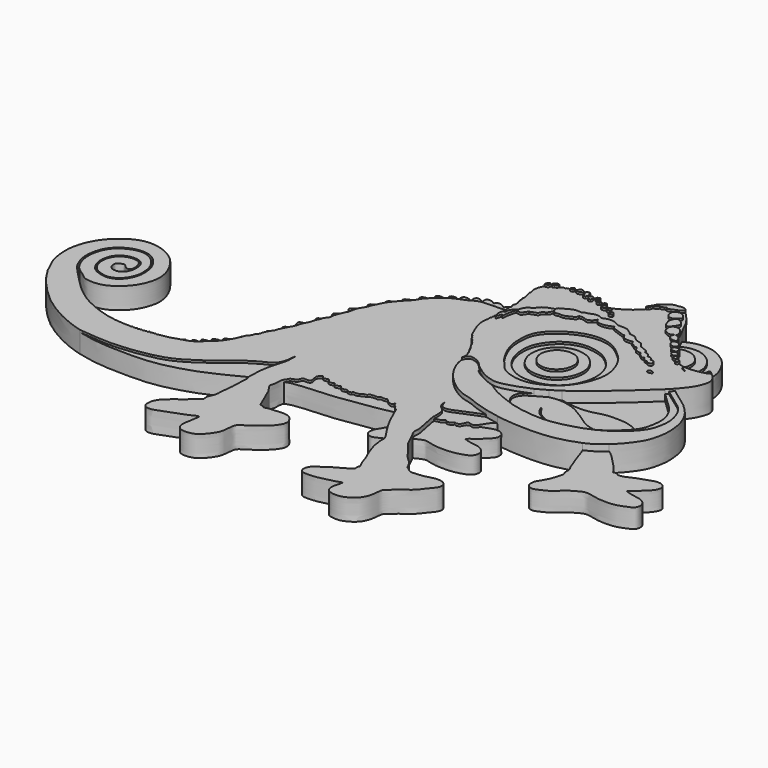
from build123d import *

# Parameters (mm, degrees)
F1_DEPTH = 4.2
F2_DEPTH = 3.9
F3_DEPTH = 3.6
F4_DEPTH = 3.3
F5_DEPTH = 3
F6_DEPTH = 2.7
F7_DEPTH = 2.4


with BuildPart() as f1:
    # F0 (on Top) → F1 (new body)
    with BuildSketch(Plane.XY):
        with BuildLine():
            add(Edge.make_bspline(
                [(4.2572836688, 14.4262746791), (4.1668524947, 14.4176068914), (3.9451777849, 14.3963399972), (3.8570355374, 13.9990727789), (3.8487542454, 13.8039519516)],
                knots=[0, 0, 0, 0, 0.1252536167, 0.3070869017, 0.3070869017, 0.3070869017, 0.3070869017], degree=3))
            add(Edge.make_bspline(
                [(3.8487542454, 13.8039519516), (3.8407848921, 13.6161809108), (3.8993235082, 13.346492022), (4.0578064985, 12.9182903306), (4.1367613559, 13.1360192483), (4.2462747554, 13.531958236), (4.3486274154, 13.7097113421), (4.395062288, 13.7903535463)],
                knots=[0.3070869017, 0.3070869017, 0.3070869017, 0.3070869017, 0.4820709135, 0.6203886142, 0.7054163793, 0.8663564139, 1, 1, 1, 1], degree=3))
            add(Edge.make_bspline(
                [(4.2572836688, 14.4262746791), (4.2510625213, 14.3391220201), (4.2456312941, 14.1150804508), (4.3258946646, 13.9316136962), (4.395062288, 13.7903535463)],
                knots=[0.3370095266, 0.3370095266, 0.3370095266, 0.3370095266, 0.3930157223, 0.4842191294, 0.4842191294, 0.4842191294, 0.4842191294], degree=3))
        make_face()
        with BuildLine():
            add(Edge.make_bspline(
                [(5.0444502362, 15.7873932545), (4.9336821254, 15.7074132414), (4.6948345412, 15.5349535618), (4.3078548058, 15.07327182), (4.2830819862, 14.6970838224), (4.2614528374, 14.4846809655), (4.2572836688, 14.4262746791)],
                knots=[0, 0, 0, 0, 0.0939097666, 0.2024961941, 0.2994763756, 0.3370095266, 0.3370095266, 0.3370095266, 0.3370095266], degree=3))
            add(Edge.make_bspline(
                [(4.2572836688, 14.4262746791), (4.2510625213, 14.3391220201), (4.2456312941, 14.1150804508), (4.3258946646, 13.9316136962), (4.395062288, 13.7903535463)],
                knots=[0.3370095266, 0.3370095266, 0.3370095266, 0.3370095266, 0.3930157223, 0.4842191294, 0.4842191294, 0.4842191294, 0.4842191294], degree=3))
            add(Edge.make_bspline(
                [(4.395062288, 13.7903535463), (4.4554023283, 13.6671218563), (4.6142712969, 13.3621522435), (4.6238515473, 13.9803985405), (4.6741068484, 14.3376181945), (4.8230768865, 15.0102517856), (4.9567118673, 15.413719314), (5.0266196335, 15.4563856567), (5.0488507354, 15.4699538176)],
                knots=[0.4842191294, 0.4842191294, 0.4842191294, 0.4842191294, 0.5637826157, 0.6524517644, 0.7470717654, 0.866413192, 0.957518569, 1, 1, 1, 1], degree=3))
            add(Edge.make_bspline(
                [(5.0444502362, 15.7873932545), (5.0251883545, 15.665911287), (5.0061965452, 15.5220360005), (5.0488507354, 15.4699538176)],
                knots=[0.4567388438, 0.4567388438, 0.4567388438, 0.4567388438, 0.5495799461, 0.5495799461, 0.5495799461, 0.5495799461], degree=3))
        make_face()
        with BuildLine():
            add(Edge.make_bspline(
                [(6.2281746506, 17.2114608534), (6.07589244, 17.1227940959), (5.7662327991, 16.9424910928), (5.3060260363, 16.5796108373), (5.1091793879, 16.1377109686), (5.0648816904, 15.9162515497), (5.0444502362, 15.7873932545)],
                knots=[0, 0, 0, 0, 0.1208192774, 0.2463555406, 0.3582604737, 0.4567388438, 0.4567388438, 0.4567388438, 0.4567388438], degree=3))
            add(Edge.make_bspline(
                [(5.0444502362, 15.7873932545), (5.0251883545, 15.665911287), (5.0061965452, 15.5220360005), (5.0488507354, 15.4699538176)],
                knots=[0.4567388438, 0.4567388438, 0.4567388438, 0.4567388438, 0.5495799461, 0.5495799461, 0.5495799461, 0.5495799461], degree=3))
            add(Edge.make_bspline(
                [(5.0488507354, 15.4699538176), (5.0819977391, 15.4294802251), (5.250436266, 15.4652867763), (5.6274792402, 15.346780719), (5.8174795469, 15.519755139), (6.1623588146, 15.9951996901), (6.1958972447, 16.1320957615), (6.2369756489, 16.1665580124)],
                knots=[0.5495799461, 0.5495799461, 0.5495799461, 0.5495799461, 0.621727708, 0.7222613953, 0.8036941472, 0.9293846552, 1, 1, 1, 1], degree=3))
            add(Edge.make_bspline(
                [(6.2281746506, 17.2114608534), (6.1135158381, 17.0160365265), (5.9480328502, 16.6862522612), (6.0321079107, 16.4493711039), (6.1503161214, 16.1992656951), (6.2369756489, 16.1665580124)],
                knots=[0.3043009144, 0.3043009144, 0.3043009144, 0.3043009144, 0.3911017829, 0.4476691528, 0.5131548523, 0.5131548523, 0.5131548523, 0.5131548523], degree=3))
        make_face()
        with BuildLine():
            add(Edge.make_bspline(
                [(8.1844923905, 18.4529813743), (7.9538408694, 18.3844008684), (7.4742727507, 18.2417556518), (6.6749524171, 17.8926337342), (6.3622454001, 17.4399708599), (6.2281746506, 17.2114608534)],
                knots=[0, 0, 0, 0, 0.0980095359, 0.2028045074, 0.3043009144, 0.3043009144, 0.3043009144, 0.3043009144], degree=3))
            add(Edge.make_bspline(
                [(6.2281746506, 17.2114608534), (6.1135158381, 17.0160365265), (5.9480328502, 16.6862522612), (6.0321079107, 16.4493711039), (6.1503161214, 16.1992656951), (6.2369756489, 16.1665580124)],
                knots=[0.3043009144, 0.3043009144, 0.3043009144, 0.3043009144, 0.3911017829, 0.4476691528, 0.5131548523, 0.5131548523, 0.5131548523, 0.5131548523], degree=3))
            add(Edge.make_bspline(
                [(6.2369756489, 16.1665580124), (6.3332888663, 16.1302067624), (6.6191498845, 16.3337159935), (7.3474795051, 16.452553548), (7.3252448852, 16.8903127533), (7.8954768308, 17.1741298045), (8.2148504477, 17.5556552492), (8.3007920074, 17.96537853), (8.2875905099, 18.1637771919)],
                knots=[0.5131548523, 0.5131548523, 0.5131548523, 0.5131548523, 0.5859355215, 0.6795756695, 0.7450454243, 0.8317172001, 0.9124531585, 1, 1, 1, 1], degree=3))
            add(Edge.make_bspline(
                [(8.1844923905, 18.4529813743), (8.2045602062, 18.3630613719), (8.246068554, 18.2649771468), (8.2875905099, 18.1637771919)],
                knots=[0.3837385117, 0.3837385117, 0.3837385117, 0.3837385117, 0.4278700646, 0.4278700646, 0.4278700646, 0.4278700646], degree=3))
        make_face()
        with BuildLine():
            add(Edge.make_bspline(
                [(10.963008211, 19.6024312746), (10.5673448659, 19.6306744746), (9.7827905716, 19.6866774482), (8.8935310005, 19.0463629809), (8.1627371569, 18.7903124531), (8.1669793995, 18.5314537016), (8.1844923905, 18.4529813743)],
                knots=[0, 0, 0, 0, 0.1239414184, 0.2457613858, 0.345225327, 0.3837385117, 0.3837385117, 0.3837385117, 0.3837385117], degree=3))
            add(Edge.make_bspline(
                [(8.1844923905, 18.4529813743), (8.2045602062, 18.3630613719), (8.246068554, 18.2649771468), (8.2875905099, 18.1637771919)],
                knots=[0.3837385117, 0.3837385117, 0.3837385117, 0.3837385117, 0.4278700646, 0.4278700646, 0.4278700646, 0.4278700646], degree=3))
            add(Edge.make_bspline(
                [(8.2875905099, 18.1637771919), (8.3688787643, 17.9656562826), (8.5328525533, 17.5421923079), (9.1945108282, 17.8529947278), (9.7420229954, 17.6601348263), (10.4929173366, 18.0831815254), (11.0825370966, 18.2972193272), (11.239049864, 18.5828948952), (11.2167243909, 18.7323113309), (11.2063457073, 18.8017721615)],
                knots=[0.4278700646, 0.4278700646, 0.4278700646, 0.4278700646, 0.5142671722, 0.6020376296, 0.6884748838, 0.7942925802, 0.8859118537, 0.9469626124, 1, 1, 1, 1], degree=3))
            add(Edge.make_bspline(
                [(10.963008211, 19.6024312746), (10.8695937544, 19.3862200958), (11.0076907657, 18.9239427064), (11.2063457073, 18.8017721615)],
                knots=[0.3861723191, 0.3861723191, 0.3861723191, 0.3861723191, 0.4955558503, 0.4955558503, 0.4955558503, 0.4955558503], degree=3))
        make_face()
        with BuildLine():
            add(Edge.make_bspline(
                [(13.4589920457, 19.857621768), (13.3678943645, 19.9353063697), (13.1528452898, 20.1186963828), (12.4045567887, 20.2592001087), (11.6220214954, 19.7919164102), (11.0452651862, 19.7928180542), (10.963008211, 19.6024312746)],
                knots=[0, 0, 0, 0, 0.0739996162, 0.173951838, 0.2898536256, 0.3861723191, 0.3861723191, 0.3861723191, 0.3861723191], degree=3))
            add(Edge.make_bspline(
                [(10.963008211, 19.6024312746), (10.8695937544, 19.3862200958), (11.0076907657, 18.9239427064), (11.2063457073, 18.8017721615)],
                knots=[0.3861723191, 0.3861723191, 0.3861723191, 0.3861723191, 0.4955558503, 0.4955558503, 0.4955558503, 0.4955558503], degree=3))
            add(Edge.make_bspline(
                [(11.2063457073, 18.8017721615), (11.3503710713, 18.7131981897), (11.6608351855, 18.8724339627), (11.8855437213, 18.7429971449), (12.4871555359, 18.5075482632), (12.8563782698, 18.7586325906), (13.1655763758, 19.0022047633), (13.3389706403, 19.2695306355), (13.3751472552, 19.3952151311), (13.3797840468, 19.4659798076)],
                knots=[0.4955558503, 0.4955558503, 0.4955558503, 0.4955558503, 0.574859203, 0.6355612787, 0.7278717029, 0.8054969368, 0.8808907464, 0.9469329265, 1, 1, 1, 1], degree=3))
            add(Edge.make_bspline(
                [(13.4589920457, 19.857621768), (13.393113852, 19.7676595789), (13.3608028601, 19.6186999468), (13.3797840468, 19.4659798076)],
                knots=[0.4575460319, 0.4575460319, 0.4575460319, 0.4575460319, 0.5375683353, 0.5375683353, 0.5375683353, 0.5375683353], degree=3))
        make_face()
        with BuildLine():
            add(Edge.make_bspline(
                [(15.9584548632, 19.6948057642), (15.7785688802, 19.7775055943), (15.4321536195, 19.9367647134), (15.0050453387, 20.2039344481), (14.2768662751, 20.2177155843), (13.7086704729, 20.0168103659), (13.5142183119, 19.9330378584), (13.4589920457, 19.857621768)],
                knots=[0, 0, 0, 0, 0.0961333952, 0.1851287945, 0.2920401615, 0.3904626346, 0.4575460319, 0.4575460319, 0.4575460319, 0.4575460319], degree=3))
            add(Edge.make_bspline(
                [(13.4589920457, 19.857621768), (13.393113852, 19.7676595789), (13.3608028601, 19.6186999468), (13.3797840468, 19.4659798076)],
                knots=[0.4575460319, 0.4575460319, 0.4575460319, 0.4575460319, 0.5375683353, 0.5375683353, 0.5375683353, 0.5375683353], degree=3))
            add(Edge.make_bspline(
                [(13.3797840468, 19.4659798076), (13.4021673605, 19.2858866014), (13.604926317, 18.8849076756), (14.3979519168, 18.7434852561), (15.2581512712, 18.9304439708), (15.7257050072, 19.188941068), (15.8433044171, 19.1953524132), (15.8836468705, 19.1975518238)],
                knots=[0.5375683353, 0.5375683353, 0.5375683353, 0.5375683353, 0.6319335793, 0.7417446274, 0.8628251639, 0.9529422007, 1, 1, 1, 1], degree=3))
            add(Edge.make_bspline(
                [(15.9584548632, 19.6948057642), (15.8750063581, 19.6546253109), (15.7393211889, 19.4733535309), (15.8636210416, 19.284672626), (15.8836468705, 19.1975518238)],
                knots=[0.422022284, 0.422022284, 0.422022284, 0.422022284, 0.4846452335, 0.5495299236, 0.5495299236, 0.5495299236, 0.5495299236], degree=3))
        make_face()
        with BuildLine():
            add(Edge.make_bspline(
                [(18.2290936964, 18.8895198406), (18.2096192844, 18.9484320287), (18.1577144311, 19.1054497854), (17.6353734729, 19.4002310133), (17.2400010001, 19.7456677316), (16.3726421884, 19.6848128688), (16.0609576479, 19.7441608527), (15.9584548632, 19.6948057642)],
                knots=[0, 0, 0, 0, 0.0546785272, 0.1457338447, 0.2345164545, 0.3451002745, 0.422022284, 0.422022284, 0.422022284, 0.422022284], degree=3))
            add(Edge.make_bspline(
                [(15.9584548632, 19.6948057642), (15.8750063581, 19.6546253109), (15.7393211889, 19.4733535309), (15.8636210416, 19.284672626), (15.8836468705, 19.1975518238)],
                knots=[0.422022284, 0.422022284, 0.422022284, 0.422022284, 0.4846452335, 0.5495299236, 0.5495299236, 0.5495299236, 0.5495299236], degree=3))
            add(Edge.make_bspline(
                [(15.8836468705, 19.1975518238), (15.9004854928, 19.1242967142), (15.8626282567, 18.939561019), (16.5551252832, 18.7459843306), (17.1614974855, 18.486365118), (17.6237553604, 18.3270215578), (17.8910943006, 18.2304738599), (17.9585837317, 18.3777258413), (17.9914677276, 18.4494738685)],
                knots=[0.5495299236, 0.5495299236, 0.5495299236, 0.5495299236, 0.6040879047, 0.7000328189, 0.8029722412, 0.8876772714, 0.9452711325, 1, 1, 1, 1], degree=3))
            add(Edge.make_bspline(
                [(18.2290936964, 18.8895198406), (18.1381372702, 18.8233146249), (18.0309103185, 18.5943745966), (17.9914677276, 18.4494738685)],
                knots=[0.3806407258, 0.3806407258, 0.3806407258, 0.3806407258, 0.4847779558, 0.4847779558, 0.4847779558, 0.4847779558], degree=3))
        make_face()
        with BuildLine():
            add(Edge.make_bspline(
                [(19.7439935147, 18.2001724016), (19.6137493842, 18.2991366797), (19.3579137313, 18.4935300127), (19.0763003482, 18.8580069705), (18.42541823, 18.870107683), (18.2856958911, 18.9307193541), (18.2290936964, 18.8895198406)],
                knots=[0, 0, 0, 0, 0.1021355922, 0.2006324663, 0.3158361153, 0.3806407258, 0.3806407258, 0.3806407258, 0.3806407258], degree=3))
            add(Edge.make_bspline(
                [(18.2290936964, 18.8895198406), (18.1381372702, 18.8233146249), (18.0309103185, 18.5943745966), (17.9914677276, 18.4494738685)],
                knots=[0.3806407258, 0.3806407258, 0.3806407258, 0.3806407258, 0.4847779558, 0.4847779558, 0.4847779558, 0.4847779558], degree=3))
            add(Edge.make_bspline(
                [(17.9914677276, 18.4494738685), (17.9635849208, 18.3470404608), (17.9783958785, 18.1976457889), (18.3266673055, 17.7086174138), (18.8570585685, 17.6334178539), (19.2473256363, 17.6342555319), (19.532957347, 17.6397288217), (19.6218028642, 17.7085537895), (19.6597432148, 17.7379021837)],
                knots=[0.4847779558, 0.4847779558, 0.4847779558, 0.4847779558, 0.5583947794, 0.66675554, 0.7734813991, 0.8666773339, 0.9431548843, 1, 1, 1, 1], degree=3))
            add(Edge.make_bspline(
                [(19.7439935147, 18.2001724016), (19.6778632235, 18.1642434182), (19.6271122968, 17.9263020006), (19.6497144289, 17.7774232499), (19.6597432148, 17.7379021837)],
                knots=[0.4335620615, 0.4335620615, 0.4335620615, 0.4335620615, 0.5200765178, 0.5548630424, 0.5548630424, 0.5548630424, 0.5548630424], degree=3))
        make_face()
        with BuildLine():
            add(Edge.make_bspline(
                [(21.1830735953, 17.2542144762), (21.1355891691, 17.3153742265), (21.0277015794, 17.4543330093), (20.7259512784, 17.7555491726), (20.6442338629, 17.9918368827), (20.0158843632, 18.0362263396), (19.8051393494, 18.2333933), (19.7439935147, 18.2001724016)],
                knots=[0, 0, 0, 0, 0.0745512869, 0.1693851925, 0.2392018667, 0.3535684829, 0.4335620615, 0.4335620615, 0.4335620615, 0.4335620615], degree=3))
            add(Edge.make_bspline(
                [(19.7439935147, 18.2001724016), (19.6778632235, 18.1642434182), (19.6271122968, 17.9263020006), (19.6497144289, 17.7774232499), (19.6597432148, 17.7379021837)],
                knots=[0.4335620615, 0.4335620615, 0.4335620615, 0.4335620615, 0.5200765178, 0.5548630424, 0.5548630424, 0.5548630424, 0.5548630424], degree=3))
            add(Edge.make_bspline(
                [(19.6597432148, 17.7379021837), (19.6722054286, 17.6887915547), (19.7249150029, 17.5588955774), (19.8314987459, 17.2755913862), (20.3229400741, 17.0982602627), (20.4248925179, 16.8348868685), (20.7311074384, 16.8409348385), (20.8522970882, 16.9047162132), (20.9091529996, 16.9346391332)],
                knots=[0.5548630424, 0.5548630424, 0.5548630424, 0.5548630424, 0.5980903202, 0.6818739731, 0.785024218, 0.8585017472, 0.933616343, 1, 1, 1, 1], degree=3))
            add(Edge.make_bspline(
                [(21.1830735953, 17.2542144762), (21.059835611, 17.2239525802), (20.9502277429, 17.0571754013), (20.9091529996, 16.9346391332)],
                knots=[0.3905667751, 0.3905667751, 0.3905667751, 0.3905667751, 0.4988002208, 0.4988002208, 0.4988002208, 0.4988002208], degree=3))
        make_face()
        with BuildLine():
            add(Edge.make_bspline(
                [(22.3129995037, 16.500930866), (22.2571519104, 16.6384700195), (22.1726570741, 16.846560424), (22.1472300401, 16.9755104232), (21.6170652768, 17.0302359179), (21.3171618568, 17.2871407291), (21.1830735953, 17.2542144762)],
                knots=[0, 0, 0, 0, 0.1027582559, 0.1554685084, 0.2728041009, 0.3905667751, 0.3905667751, 0.3905667751, 0.3905667751], degree=3))
            add(Edge.make_bspline(
                [(21.1830735953, 17.2542144762), (21.059835611, 17.2239525802), (20.9502277429, 17.0571754013), (20.9091529996, 16.9346391332)],
                knots=[0.3905667751, 0.3905667751, 0.3905667751, 0.3905667751, 0.4988002208, 0.4988002208, 0.4988002208, 0.4988002208], degree=3))
            add(Edge.make_bspline(
                [(20.9091529996, 16.9346391332), (20.8808349937, 16.8501594144), (20.8894120755, 16.7222970837), (21.0961061557, 16.5992709533), (21.0813896287, 16.3171855552), (21.504250895, 16.217662597), (21.7755730437, 16.0808493651), (21.9012105239, 16.1886698722), (21.9591845792, 16.238422478)],
                knots=[0.4988002208, 0.4988002208, 0.4988002208, 0.4988002208, 0.5734191984, 0.6491660272, 0.7284327536, 0.8333863433, 0.9231179316, 1, 1, 1, 1], degree=3))
            add(Edge.make_bspline(
                [(22.3129995037, 16.500930866), (22.2194654968, 16.4797428909), (22.1009697173, 16.3629083803), (21.968345462, 16.2884854551), (21.9591845792, 16.238422478)],
                knots=[0.3362843473, 0.3362843473, 0.3362843473, 0.3362843473, 0.430913951, 0.5081963418, 0.5081963418, 0.5081963418, 0.5081963418], degree=3))
        make_face()
        with BuildLine():
            add(Edge.make_bspline(
                [(23.1467128984, 15.8916513105), (23.1099803769, 16.0054034322), (23.0359728991, 16.2345874707), (22.7406811556, 16.4485436094), (22.4299309185, 16.527418985), (22.3129995037, 16.500930866)],
                knots=[0, 0, 0, 0, 0.1081927869, 0.2179832734, 0.3362843473, 0.3362843473, 0.3362843473, 0.3362843473], degree=3))
            add(Edge.make_bspline(
                [(22.3129995037, 16.500930866), (22.2194654968, 16.4797428909), (22.1009697173, 16.3629083803), (21.968345462, 16.2884854551), (21.9591845792, 16.238422478)],
                knots=[0.3362843473, 0.3362843473, 0.3362843473, 0.3362843473, 0.430913951, 0.5081963418, 0.5081963418, 0.5081963418, 0.5081963418], degree=3))
            add(Edge.make_bspline(
                [(21.9591845792, 16.238422478), (21.9484207184, 16.1795994443), (22.0769337463, 16.0012313233), (22.2456058944, 15.7208014323), (22.561113977, 15.5394749048), (22.8258299171, 15.3691560668), (22.9565100815, 15.4753858265), (23.0177696445, 15.5251836567)],
                knots=[0.5081963418, 0.5081963418, 0.5081963418, 0.5081963418, 0.5990016623, 0.7063231478, 0.8177154214, 0.9145495901, 1, 1, 1, 1], degree=3))
            add(Edge.make_bspline(
                [(23.1467128984, 15.8916513105), (23.0721241144, 15.8310132467), (23.0028122965, 15.6833543329), (22.997325434, 15.5763155101), (23.0177696445, 15.5251836567)],
                knots=[0.3952835807, 0.3952835807, 0.3952835807, 0.3952835807, 0.5116622834, 0.6023690655, 0.6023690655, 0.6023690655, 0.6023690655], degree=3))
        make_face()
        with BuildLine():
            add(Edge.make_bspline(
                [(23.9076043184, 15.5242508002), (23.8635907958, 15.5984029745), (23.7649479764, 15.7494575978), (23.5090385532, 16.044027998), (23.2342977745, 15.9628547411), (23.1467128984, 15.8916513105)],
                knots=[0, 0, 0, 0, 0.1206748225, 0.2586274549, 0.3952835807, 0.3952835807, 0.3952835807, 0.3952835807], degree=3))
            add(Edge.make_bspline(
                [(23.1467128984, 15.8916513105), (23.0721241144, 15.8310132467), (23.0028122965, 15.6833543329), (22.997325434, 15.5763155101), (23.0177696445, 15.5251836567)],
                knots=[0.3952835807, 0.3952835807, 0.3952835807, 0.3952835807, 0.5116622834, 0.6023690655, 0.6023690655, 0.6023690655, 0.6023690655], degree=3))
            add(Edge.make_bspline(
                [(23.0177696445, 15.5251836567), (23.0470837573, 15.4518677944), (23.2109390254, 15.2756404276), (23.5180032713, 14.9579423124), (23.7072306659, 15.0306915663), (23.7924764131, 15.066357291)],
                knots=[0.6023690655, 0.6023690655, 0.6023690655, 0.6023690655, 0.7324297908, 0.8817217829, 1, 1, 1, 1], degree=3))
            add(Edge.make_bspline(
                [(23.9076043184, 15.5242508002), (23.8520162254, 15.4832744487), (23.8247358937, 15.3202437291), (23.776657275, 15.1468849053), (23.7924764131, 15.066357291)],
                knots=[0.5956140984, 0.5956140984, 0.5956140984, 0.5956140984, 0.6967312905, 0.8076016597, 0.8076016597, 0.8076016597, 0.8076016597], degree=3))
        make_face()
        with BuildLine():
            add(Edge.make_bspline(
                [(24.0698286585, 14.8099381092), (24.1413414433, 14.7917967532), (24.3122164688, 14.7696490247), (24.5909874328, 14.9108880866), (24.5166655814, 15.3159289855), (24.2329320084, 15.5674267848), (23.9722453644, 15.571900469), (23.9076043184, 15.5242508002)],
                knots=[0, 0, 0, 0, 0.1066298334, 0.216703929, 0.3447999093, 0.4780291857, 0.5956140984, 0.5956140984, 0.5956140984, 0.5956140984], degree=3))
            add(Edge.make_bspline(
                [(23.9076043184, 15.5242508002), (23.8520162254, 15.4832744487), (23.8247358937, 15.3202437291), (23.776657275, 15.1468849053), (23.7924764131, 15.066357291)],
                knots=[0.5956140984, 0.5956140984, 0.5956140984, 0.5956140984, 0.6967312905, 0.8076016597, 0.8076016597, 0.8076016597, 0.8076016597], degree=3))
            add(Edge.make_bspline(
                [(23.7924764131, 15.066357291), (23.8068148699, 14.9933671117), (23.8987001614, 14.8695729151), (24.0081909486, 14.8255743571), (24.0698286585, 14.8099381092)],
                knots=[0.8076016597, 0.8076016597, 0.8076016597, 0.8076016597, 0.908094493, 1, 1, 1, 1], degree=3))
        make_face()
    extrude(amount=F1_DEPTH)



with BuildPart() as f1b:
    # F0 (on Top) → F1, piece 2 (new body)
    with BuildSketch(Plane.XY):
        with BuildLine():
            add(Edge.make_bspline(
                [(3.5371385055, 22.3215147468), (3.5457901494, 22.3356327377), (3.4509671779, 22.4523634942), (3.5799017954, 22.7321377655), (3.8995714106, 22.9626252171), (4.0582481608, 22.8256596666), (4.0966159972, 22.8158241739)],
                knots=[0.0415505514, 0.0415505514, 0.0415505514, 0.0415505514, 0.0440912282, 0.0481156422, 0.0525177879, 0.0557967633, 0.0557967633, 0.0557967633, 0.0557967633], degree=3))
            add(Edge.make_bspline(
                [(3.5371385055, 22.3215147468), (3.6271019702, 22.2823788674), (3.743740294, 22.3842223081), (4.0245600236, 22.3241812683), (3.9918292835, 22.6585635122), (4.1190064241, 22.7494917217), (4.0966159972, 22.8158241739)],
                knots=[0, 0, 0, 0, 0.2545794284, 0.4968595849, 0.7679540305, 1, 1, 1, 1], degree=3))
        make_face()
    extrude(amount=F1_DEPTH)


with BuildPart() as f1c:
    # F0 (on Top) → F1, piece 3 (new body)
    with BuildSketch(Plane.XY):
        with BuildLine():
            add(Edge.make_bspline(
                [(4.1312665384, 22.8306749341), (4.1473100978, 22.8644015969), (4.1245228601, 23.0817393587), (4.5806274605, 23.4289458454), (4.8460903908, 23.2414101542), (4.9034759929, 23.2266794286)],
                knots=[0.0572288676, 0.0572288676, 0.0572288676, 0.0572288676, 0.0606386556, 0.0658671601, 0.0700460145, 0.0700460145, 0.0700460145, 0.0700460145], degree=3))
            add(Edge.make_bspline(
                [(4.9034759929, 23.2266794286), (4.887991338, 23.1627901912), (4.8608529788, 23.0470164804), (4.8461884631, 22.791323541), (4.6396048732, 22.9668492453), (4.5423498251, 22.7228472594), (4.3902895848, 22.7789681125), (4.3026578415, 22.6634020729), (4.1922227387, 22.7734570634), (4.1312665384, 22.8306749341)],
                knots=[0, 0, 0, 0, 0.1596795631, 0.3067673369, 0.4457574827, 0.5993737568, 0.7256156151, 0.8373430366, 1, 1, 1, 1], degree=3))
        make_face()
    extrude(amount=F1_DEPTH)


with BuildPart() as f1d:
    # F0 (on Top) → F1, piece 4 (new body)
    with BuildSketch(Plane.XY):
        with BuildLine():
            add(Edge.make_bspline(
                [(7.4280085898, 23.8107856636), (7.4377306283, 23.8092717106), (7.5052841257, 23.8945318365), (7.7727009058, 23.7995672352), (7.8282719507, 23.756057801), (7.8537141116, 23.7662353551)],
                knots=[0.1156454597, 0.1156454597, 0.1156454597, 0.1156454597, 0.1177851056, 0.1216447401, 0.1238292275, 0.1238292275, 0.1238292275, 0.1238292275], degree=3))
            add(Edge.make_bspline(
                [(7.4280085898, 23.8107856636), (7.3766564638, 23.7475123489), (7.2735661525, 23.6204900382), (7.0566038195, 23.3666938131), (7.4035654765, 23.1331394567), (7.8593625318, 23.361660571), (8.1399858659, 23.4493261795), (7.9929646677, 23.6574600269), (7.9002610526, 23.7298752936), (7.8537141116, 23.7662353551)],
                knots=[0, 0, 0, 0, 0.1405204316, 0.2820972792, 0.4303513066, 0.6303391904, 0.7614221214, 0.8802088739, 1, 1, 1, 1], degree=3))
        make_face()
    extrude(amount=F1_DEPTH)


with BuildPart() as f1e:
    # F0 (on Top) → F1, piece 5 (new body)
    with BuildSketch(Plane.XY):
        with BuildLine():
            add(Edge.make_bspline(
                [(8.3685202503, 23.7711856086), (8.4411550274, 23.7767863775), (8.6048472617, 23.9564383883), (8.7853257036, 23.728075442), (8.8585766011, 23.7068342865)],
                knots=[0.1347926544, 0.1347926544, 0.1347926544, 0.1347926544, 0.1384613677, 0.142482163, 0.142482163, 0.142482163, 0.142482163], degree=3))
            add(Edge.make_bspline(
                [(8.3685202503, 23.7711856086), (8.3089620328, 23.7163065337), (8.1969474117, 23.6130922497), (8.2457773916, 23.4039641918), (8.3902356318, 23.3308379705), (8.46887727, 23.2910287784)],
                knots=[0, 0, 0, 0, 0.3409313668, 0.6412095501, 1, 1, 1, 1], degree=3))
            add(Edge.make_bspline(
                [(8.46887727, 23.2910287784), (8.5210476686, 23.3929454982), (8.6708410978, 23.5104995137), (8.7956695287, 23.534663096), (8.8554762831, 23.5043294781)],
                knots=[0.5758086521, 0.5758086521, 0.5758086521, 0.5758086521, 0.7247932359, 0.8385048543, 0.8385048543, 0.8385048543, 0.8385048543], degree=3))
            add(Edge.make_bspline(
                [(8.8585766011, 23.7068342865), (8.882666562, 23.6660600925), (8.9280929014, 23.5891723637), (8.8786834817, 23.5314440112), (8.8554762831, 23.5043294781)],
                knots=[0, 0, 0, 0, 0.5303082127, 1, 1, 1, 1], degree=3))
        make_face()
        with BuildLine():
            add(Edge.make_bspline(
                [(8.46887727, 23.2910287784), (8.5210476686, 23.3929454982), (8.6708410978, 23.5104995137), (8.7956695287, 23.534663096), (8.8554762831, 23.5043294781)],
                knots=[0.5758086521, 0.5758086521, 0.5758086521, 0.5758086521, 0.7247932359, 0.8385048543, 0.8385048543, 0.8385048543, 0.8385048543], degree=3))
            add(Edge.make_bspline(
                [(9.0325375779, 23.2042514279), (9.0277179376, 23.062005779), (8.8280647343, 22.8188321366), (8.6623791576, 22.8408557448), (8.379611749, 22.9072554718), (8.412760722, 23.181403116), (8.46887727, 23.2910287784)],
                knots=[0, 0, 0, 0, 0.1745100693, 0.2837135416, 0.4155549302, 0.5758086521, 0.5758086521, 0.5758086521, 0.5758086521], degree=3))
            add(Edge.make_bspline(
                [(8.8554762831, 23.5043294781), (8.9404148376, 23.4612491657), (9.0369977704, 23.3358884268), (9.0325375779, 23.2042514279)],
                knots=[0.8385048543, 0.8385048543, 0.8385048543, 0.8385048543, 1, 1, 1, 1], degree=3))
        make_face()
    extrude(amount=F1_DEPTH)


with BuildPart() as f1f:
    # F0 (on Top) → F1, piece 6 (new body)
    with BuildSketch(Plane.XY):
        with BuildLine():
            add(Edge.make_bspline(
                [(10.0614418309, 23.4296319293), (10.1264019942, 23.4512446083), (10.2818185649, 23.5644330528), (10.4973149991, 23.5549430821), (10.5737897551, 23.3272905166), (10.6108992504, 23.2910287784)],
                knots=[0.1626365822, 0.1626365822, 0.1626365822, 0.1626365822, 0.166342194, 0.1695193261, 0.1732669684, 0.1732669684, 0.1732669684, 0.1732669684], degree=3))
            add(Edge.make_bspline(
                [(10.6108992504, 23.2910287784), (10.6174624982, 23.2592490484), (10.6328955454, 23.1845210963), (10.4705985624, 23.086300132), (10.2110122618, 23.0067329351), (10.0015830348, 23.1006747089), (9.9865094104, 23.2971658348), (10.0369600108, 23.3863527842), (10.0614418309, 23.4296319293)],
                knots=[0, 0, 0, 0, 0.122196948, 0.2873381133, 0.4991002904, 0.6777481908, 0.8436230539, 1, 1, 1, 1], degree=3))
        make_face()
    extrude(amount=F1_DEPTH)


with BuildPart() as f1g:
    # F0 (on Top) → F1, piece 7 (new body)
    with BuildSketch(Plane.XY):
        with BuildLine():
            add(Edge.make_bspline(
                [(11.5469813216, 22.934095786), (11.5870790982, 22.9460737153), (11.7669108618, 23.0309884794), (11.9377295408, 22.8537877141), (11.9626729753, 22.7466490423), (11.9814410018, 22.7329419431)],
                knots=[0.1843385395, 0.1843385395, 0.1843385395, 0.1843385395, 0.1876997953, 0.1912022887, 0.19373915, 0.19373915, 0.19373915, 0.19373915], degree=3))
            add(Edge.make_bspline(
                [(11.5469813216, 22.934095786), (11.5179383135, 22.9012428002), (11.4577019915, 22.8331044373), (11.326053844, 22.7007027433), (11.4580983344, 22.506215938), (11.6014402264, 22.4591401386), (11.7996152484, 22.5367787405), (11.9666129346, 22.6709221003), (11.977672995, 22.7171818857), (11.9814410018, 22.7329419431)],
                knots=[0, 0, 0, 0, 0.1355780298, 0.2811940769, 0.4424816267, 0.5792231955, 0.7472362242, 0.9138869412, 1, 1, 1, 1], degree=3))
        make_face()
    extrude(amount=F1_DEPTH)


with BuildPart() as f1h:
    # F0 (on Top) → F1, piece 8 (new body)
    with BuildSketch(Plane.XY):
        with BuildLine():
            add(Edge.make_bspline(
                [(26.5533431796, 17.2253629794), (26.5647290162, 17.1522633622), (26.5867506747, 17.0108793894), (26.4157431674, 16.8773824015), (26.0891959114, 16.9543457507), (26.0385711479, 17.2219582086), (26.0356002192, 17.3643092541), (26.1821467116, 17.4283796529), (26.267794419, 17.4658249898)],
                knots=[0, 0, 0, 0, 0.1644412435, 0.3180503154, 0.5142854773, 0.6950628088, 0.8217823511, 1, 1, 1, 1], degree=3))
            add(Edge.make_bspline(
                [(26.5533431796, 17.2253629794), (26.5216691995, 17.2685313543), (26.5002147076, 17.3757232088), (26.3553995993, 17.4089749987), (26.2918422104, 17.4407928506), (26.267794419, 17.4658249898)],
                knots=[0.7851609802, 0.7851609802, 0.7851609802, 0.7851609802, 0.8436714648, 0.8984560026, 0.9470322164, 0.9470322164, 0.9470322164, 0.9470322164], degree=3))
        make_face()
    extrude(amount=F1_DEPTH)


with BuildPart() as f1i:
    # F0 (on Top) → F1, piece 9 (new body)
    with BuildSketch(Plane.XY):
        with BuildLine():
            add(Edge.make_bspline(
                [(15.611296156, 25.104438738), (15.64030298, 25.1751928819), (15.5785250356, 25.3006500907), (15.9927159955, 25.7385654654), (16.0231873238, 25.7436582677), (16.0302138154, 25.7579214924)],
                knots=[0.2250532894, 0.2250532894, 0.2250532894, 0.2250532894, 0.2284059472, 0.2338385821, 0.2354167121, 0.2354167121, 0.2354167121, 0.2354167121], degree=3))
            add(Edge.make_bspline(
                [(15.611296156, 25.104438738), (15.6179964797, 25.0777863179), (15.639017182, 24.9941705681), (15.9973038919, 25.1911159485), (16.0214482437, 25.4568116466), (16.0673150307, 25.6098758229), (16.0894018851, 25.6835828863)],
                knots=[0, 0, 0, 0, 0.1453725026, 0.4560723099, 0.7380751417, 1, 1, 1, 1], degree=3))
            add(Edge.make_bspline(
                [(16.0302138154, 25.7579214924), (16.0430171637, 25.7238166214), (16.0558233133, 25.689712793), (16.0894018851, 25.6835828863)],
                knots=[0, 0, 0, 0, 0.1637534305, 0.1637534305, 0.1637534305, 0.1637534305], degree=3))
        make_face()
        with BuildLine():
            add(Edge.make_bspline(
                [(17.5397924016, 26.4365977838), (17.5299817617, 26.3184081346), (17.5719321739, 26.1195787023), (17.7999932306, 26.1846061715), (18.6522474071, 26.5514648806), (19.3371308864, 26.8218667037), (19.5153950838, 27.0134254278), (19.5863430916, 27.0896464326)],
                knots=[0.3257562689, 0.3257562689, 0.3257562689, 0.3257562689, 0.4219799438, 0.5052871654, 0.7037292406, 0.8821455065, 1, 1, 1, 1], degree=3))
            add(Edge.make_bspline(
                [(18.2136354947, 27.389219321), (18.2713229309, 27.3875399756), (18.5101256085, 27.5405709368), (19.0540359725, 27.4493308911), (19.3574624457, 27.4202284245), (19.5249055621, 27.1808069188), (19.5863430916, 27.0896464326)],
                knots=[0.2701484653, 0.2701484653, 0.2701484653, 0.2701484653, 0.2741688072, 0.2796394935, 0.284144628, 0.2868747246, 0.2868747246, 0.2868747246, 0.2868747246], degree=3))
            add(Edge.make_bspline(
                [(18.2136354947, 27.389219321), (18.1121141506, 27.2977925186), (17.8879034408, 27.0958757074), (17.5805923186, 26.7118227063), (17.5426270043, 26.4707464936), (17.5397924016, 26.4365977838)],
                knots=[0, 0, 0, 0, 0.1349074957, 0.2979542206, 0.3257562689, 0.3257562689, 0.3257562689, 0.3257562689], degree=3))
        make_face()
        with BuildLine():
            add(Edge.make_bspline(
                [(16.0302138154, 25.7579214924), (16.0472807107, 25.792565946), (16.0887750321, 26.0500455547), (16.3353610072, 26.4265822623), (16.6149151643, 26.5537224526), (16.8972602269, 26.7194636674), (17.0465439666, 26.8613343717), (17.0799175461, 26.8942939464)],
                knots=[0.2354167121, 0.2354167121, 0.2354167121, 0.2354167121, 0.2392498882, 0.2442265228, 0.2482787503, 0.253161828, 0.2545908019, 0.2545908019, 0.2545908019, 0.2545908019], degree=3))
            add(Edge.make_bspline(
                [(16.0302138154, 25.7579214924), (16.0430171637, 25.7238166214), (16.0558233133, 25.689712793), (16.0894018851, 25.6835828863)],
                knots=[0, 0, 0, 0, 0.1637534305, 0.1637534305, 0.1637534305, 0.1637534305], degree=3))
            add(Edge.make_bspline(
                [(16.0894018851, 25.6835828863), (16.1522075901, 25.6721174459), (16.4147843914, 25.8395743481), (16.6122413803, 25.9528364441), (16.7250869345, 26.140078887), (16.7281423645, 26.1397474107)],
                knots=[0.1637534305, 0.1637534305, 0.1637534305, 0.1637534305, 0.4700395261, 0.7573879409, 0.9793998437, 0.9793998437, 0.9793998437, 0.9793998437], degree=3))
            add(Edge.make_bspline(
                [(17.0799175461, 26.8942939464), (16.9348348417, 26.6255942557), (16.7627869406, 26.3079773044), (16.727979369, 26.1583335254), (16.7281423645, 26.1397474107)],
                knots=[0, 0, 0, 0, 0.3454837227, 0.4088575218, 0.4088575218, 0.4088575218, 0.4088575218], degree=3))
        make_face()
        with BuildLine():
            add(Edge.make_bspline(
                [(18.2136354947, 27.389219321), (18.1121141506, 27.2977925186), (17.8879034408, 27.0958757074), (17.5805923186, 26.7118227063), (17.5426270043, 26.4707464936), (17.5397924016, 26.4365977838)],
                knots=[0, 0, 0, 0, 0.1349074957, 0.2979542206, 0.3257562689, 0.3257562689, 0.3257562689, 0.3257562689], degree=3))
            add(Edge.make_bspline(
                [(17.0799175461, 26.8942939464), (17.1712243121, 26.9844680366), (17.3761718232, 27.2087843654), (17.7711509946, 27.3835191686), (18.1276699792, 27.4526093546), (18.1814163206, 27.3901572569), (18.2136354947, 27.389219321)],
                knots=[0.2545908019, 0.2545908019, 0.2545908019, 0.2545908019, 0.2585003313, 0.2636809883, 0.2679030528, 0.2701484653, 0.2701484653, 0.2701484653, 0.2701484653], degree=3))
            add(Edge.make_bspline(
                [(17.0799175461, 26.8942939464), (16.9348348417, 26.6255942557), (16.7627869406, 26.3079773044), (16.727979369, 26.1583335254), (16.7281423645, 26.1397474107)],
                knots=[0, 0, 0, 0, 0.3454837227, 0.4088575218, 0.4088575218, 0.4088575218, 0.4088575218], degree=3))
            add(Edge.make_bspline(
                [(16.7281423645, 26.1397474107), (16.7284258733, 26.1397166535), (16.7283122171, 26.1389803845), (16.7281679757, 26.1382438256)],
                knots=[0.9793998437, 0.9793998437, 0.9793998437, 0.9793998437, 1, 1, 1, 1], degree=3))
            add(Edge.make_bspline(
                [(16.7281679757, 26.1382438256), (16.7286676626, 26.1186025116), (16.7613604523, 26.0511562692), (17.1986628646, 26.1722795375), (17.4232832831, 26.3464787936), (17.5397924016, 26.4365977838)],
                knots=[0.4105780625, 0.4105780625, 0.4105780625, 0.4105780625, 0.4784654559, 0.7299984274, 1, 1, 1, 1], degree=3))
        make_face()
    extrude(amount=F1_DEPTH)


with BuildPart() as f1j:
    # F0 (on Top) → F1, piece 10 (new body)
    with BuildSketch(Plane.XY):
        with BuildLine():
            add(Edge.make_bspline(
                [(22.922639974, 21.5966674827), (22.957692749, 21.5663303832), (23.0696935914, 21.5559172872), (23.2140521764, 21.0985789272), (23.2692898504, 21.0189176886)],
                knots=[0.1157794896, 0.1157794896, 0.1157794896, 0.1157794896, 0.1356082083, 0.1736867174, 0.1736867174, 0.1736867174, 0.1736867174], degree=3))
            add(Edge.make_bspline(
                [(23.2692898504, 21.0189176886), (23.2950655567, 20.9616436242), (23.3485516664, 20.8427990254), (23.1327365156, 20.7246811601), (22.6785811495, 20.7249096478), (22.2864174076, 21.0105713187), (22.0551608218, 21.2244375668), (22.077277789, 21.6644427543), (22.3766537299, 21.8793240748), (22.6112126976, 21.8468550335), (22.7947011413, 21.7061728977), (22.8811722337, 21.6316998935), (22.922639974, 21.5966674827)],
                knots=[0, 0, 0, 0, 0.0763916387, 0.1585617392, 0.2848984785, 0.4156133678, 0.5188284916, 0.63627407, 0.7448209372, 0.8330811305, 0.9225959717, 1, 1, 1, 1], degree=3))
        make_face()
    extrude(amount=F1_DEPTH)


with BuildPart() as f1k:
    # F0 (on Top) → F1, piece 11 (new body)
    with BuildSketch(Plane.XY):
        with BuildLine():
            add(Edge.make_bspline(
                [(25.7833942931, 17.9431058431), (25.6964929308, 17.9492330562), (25.5339369692, 17.960732767), (25.3898180883, 17.8190400657), (25.3164140679, 17.5834466874), (25.5841534476, 17.3579650707), (25.8473580378, 17.3668476223), (26.0091332257, 17.5050062353), (26.0068087259, 17.6487619585), (26.0058796254, 17.7230952221)],
                knots=[0, 0, 0, 0, 0.1482002881, 0.2773293444, 0.4156689466, 0.5821800886, 0.7327734789, 0.8621330204, 1, 1, 1, 1], degree=3))
            add(Edge.make_bspline(
                [(25.7833942931, 17.9431058431), (25.8032494779, 17.924652214), (25.8756975646, 17.8570412261), (25.9483588554, 17.7778920987), (26.0058796254, 17.7230952221)],
                knots=[0.6436691139, 0.6436691139, 0.6436691139, 0.6436691139, 0.6504795011, 0.6682048633, 0.6682048633, 0.6682048633, 0.6682048633], degree=3))
        make_face()
    extrude(amount=F1_DEPTH)


with BuildPart() as f1l:
    # F0 (on Top) → F1, piece 12 (new body)
    with BuildSketch(Plane.XY):
        with BuildLine():
            add(Edge.make_bspline(
                [(23.5389051061, 20.6401700536), (23.5806108088, 20.5808679088), (23.9585720055, 20.5773882997), (24.1302424842, 20.2202419409), (24.179087452, 19.9743306901), (24.2129462038, 19.8890963075)],
                knots=[0.253418249, 0.253418249, 0.253418249, 0.253418249, 0.2850932059, 0.3170973922, 0.3470983767, 0.3470983767, 0.3470983767, 0.3470983767], degree=3))
            add(Edge.make_bspline(
                [(24.2129462038, 19.8890963075), (24.2075313251, 19.8333148638), (24.1953232254, 19.7085526835), (23.9262284893, 19.5908412085), (23.5668316641, 19.579111682), (23.3338463298, 19.7453405086), (23.0811589799, 20.0451418132), (23.0223659605, 20.3839325732), (23.1877947416, 20.5645716815), (23.4202964375, 20.6092756737), (23.5389051061, 20.6401700536)],
                knots=[0, 0, 0, 0, 0.0938835079, 0.2147945906, 0.3532278556, 0.4761392507, 0.6223764402, 0.7531250441, 0.8600344915, 1, 1, 1, 1], degree=3))
        make_face()
    extrude(amount=F1_DEPTH)


with BuildPart() as f1m:
    # F0 (on Top) → F1, piece 13 (new body)
    with BuildSketch(Plane.XY):
        with BuildLine():
            add(Edge.make_bspline(
                [(25.1630240811, 18.656564071), (25.1227224456, 18.6647000277), (25.0254920217, 18.6843280086), (24.7485091999, 18.6614813917), (24.5394940691, 18.4587926221), (24.6835264852, 18.1602543743), (24.8737292446, 17.9448625942), (25.0864844967, 17.8955916011), (25.3203107909, 17.9393074751), (25.4440223599, 18.0641141531), (25.5308200201, 18.2059135122), (25.5049285588, 18.3297613982)],
                knots=[0, 0, 0, 0, 0.0854459136, 0.2061791327, 0.3197386617, 0.4454370738, 0.5692951862, 0.6749379681, 0.7844104409, 0.8788337291, 1, 1, 1, 1], degree=3))
            add(Edge.make_bspline(
                [(25.1630240811, 18.656564071), (25.2067372322, 18.627831241), (25.3214250281, 18.6349702224), (25.4193604342, 18.5487559948), (25.4747956475, 18.4020562878), (25.5049285588, 18.3297613982)],
                knots=[0.5460150264, 0.5460150264, 0.5460150264, 0.5460150264, 0.5662595386, 0.5860308076, 0.6041812699, 0.6041812699, 0.6041812699, 0.6041812699], degree=3))
        make_face()
    extrude(amount=F1_DEPTH)


with BuildPart() as f1n:
    # F0 (on Top) → F1, piece 14 (new body)
    with BuildSketch(Plane.XY):
        with BuildLine():
            add(Edge.make_bspline(
                [(24.4440461214, 19.5745441897), (24.4780775575, 19.5607885267), (24.5517485935, 19.5881176713), (24.6743548262, 19.4981318763), (24.8466462041, 19.462044393), (24.9295066286, 19.2116868002), (24.9114403714, 19.1107246748), (24.9255046118, 19.0609879407)],
                knots=[0.3930212753, 0.3930212753, 0.3930212753, 0.3930212753, 0.4096468646, 0.4290929153, 0.4502423234, 0.4754212983, 0.4957988573, 0.4957988573, 0.4957988573, 0.4957988573], degree=3))
            add(Edge.make_bspline(
                [(24.9255046118, 19.0609879407), (24.9216912823, 19.0142589292), (24.9126389346, 18.90333034), (24.6575249821, 18.7267289631), (24.2621742592, 18.8069850956), (23.9924953733, 18.940339937), (23.9668323968, 19.3019842861), (24.0247769762, 19.5341725474), (24.2870687827, 19.5486970895), (24.394804714, 19.5664363469), (24.4440461214, 19.5745441897)],
                knots=[0, 0, 0, 0, 0.0953984752, 0.2264635596, 0.3850363322, 0.5172567541, 0.66270267, 0.7777190427, 0.8984050442, 1, 1, 1, 1], degree=3))
        make_face()
    extrude(amount=F1_DEPTH)


with BuildPart() as f1o:
    # F0 (on Top) → F1, piece 15 (new body)
    with BuildSketch(Plane.XY):
        with BuildLine():
            add(Edge.make_bspline(
                [(21.9098082668, 23.1440910575), (21.7115719589, 23.2718392499), (21.1506115732, 23.4908672482), (20.5905425028, 23.0034155858), (20.6330800878, 22.4869648557), (20.7481437273, 22.0078784075), (21.176476421, 21.7736247471), (21.7879038707, 21.4955134346), (22.1730092799, 21.830327694), (22.5285097394, 21.9336188091), (22.4661002501, 22.2349678265), (22.2709902114, 22.8087214953), (22.0698111266, 23.0409814085), (21.9098082668, 23.1440910575)],
                knots=[0, 0, 0, 0, 0.1135191887, 0.2149119256, 0.3053482261, 0.3926598024, 0.4818898125, 0.5833430145, 0.6723894457, 0.7443155469, 0.8082169578, 0.9083750347, 1, 1, 1, 1], degree=3))
        make_face()
    extrude(amount=F1_DEPTH)


with BuildPart() as f1p:
    # F0 (on Top) → F1, piece 16 (new body)
    with BuildSketch(Plane.XY):
        with BuildLine():
            add(Edge.make_bspline(
                [(20.4440737341, 22.9761413845), (20.5688812347, 23.0597692887), (20.9417360669, 23.4247028819), (21.3384649293, 24.1770721071), (20.9600356446, 24.5648911536), (20.5446000868, 24.9319764935), (20.0818048259, 24.9911962915), (19.8197179397, 24.6756342572), (19.5920025066, 24.1784009723), (19.7271364184, 23.6711846441), (19.9368994919, 23.1236473691), (20.2575568337, 22.887813075), (20.3778593806, 22.9317741182), (20.4440737341, 22.9761413845)],
                knots=[0, 0, 0, 0, 0.1069872476, 0.2230584141, 0.3124494573, 0.4110649828, 0.4945416677, 0.574837846, 0.6699952664, 0.7647128559, 0.8661296381, 0.9432398581, 1, 1, 1, 1], degree=3))
        make_face()
    extrude(amount=F1_DEPTH)


with BuildPart() as f1q:
    # F0 (on Top) → F1, piece 17 (new body)
    with BuildSketch(Plane.XY):
        with BuildLine():
            add(Edge.make_bspline(
                [(19.3867568015, 24.7052530647), (19.5889572511, 24.7180571265), (20.0223802155, 25.0029501182), (20.6353792829, 25.4946632833), (19.9211558353, 26.1924117919), (19.4199404391, 26.347496022), (18.8425835071, 26.1682382385), (18.5371591938, 25.7006555609), (18.7246765287, 25.0767244854), (18.9586222104, 24.8298882234), (19.2298113131, 24.6953147103), (19.3867568015, 24.7052530647)],
                knots=[0, 0, 0, 0, 0.1257795168, 0.2428881654, 0.3752771709, 0.484561838, 0.5946580048, 0.7005211211, 0.8155539171, 0.9023714945, 1, 1, 1, 1], degree=3))
        make_face()
    extrude(amount=F1_DEPTH)


with BuildPart() as f1r:
    # F0 (on Top) → F1, piece 18 (new body)
    with BuildSketch(Plane.XY):
        with BuildLine():
            add(Edge.make_bspline(
                [(13.915550367, 21.2962383786), (13.8934881799, 21.2320067914), (13.6910384683, 21.172757163), (13.4718661821, 21.1078823979), (13.2399185401, 21.3979024049), (13.383095335, 21.6051542084), (13.6362117972, 21.7611043673), (13.7354662552, 21.7343171253), (13.8107724371, 21.5629257657), (13.9393385028, 21.365494872), (13.915550367, 21.2962383786)],
                knots=[0, 0, 0, 0, 0.1314450489, 0.257281717, 0.4006089236, 0.5265421133, 0.6687493863, 0.7426725681, 0.8582718635, 1, 1, 1, 1], degree=3))
        make_face()
    extrude(amount=F1_DEPTH)


with BuildPart() as f1s:
    # F0 (on Top) → F1, piece 19 (new body)
    with BuildSketch(Plane.XY):
        with BuildLine():
            add(Edge.make_bspline(
                [(12.8316835096, 21.8047694302), (12.9324325074, 21.79566528), (13.1126770368, 21.8115756194), (13.1829018018, 21.9329171921), (13.1455403477, 22.1697162444), (12.9510038076, 22.3224283273), (12.8029094651, 22.3233433292), (12.5227985424, 22.162628557), (12.5623527351, 21.99412116), (12.5892350548, 21.8557547502), (12.7380163777, 21.8132336299), (12.8316835096, 21.8047694302)],
                knots=[0, 0, 0, 0, 0.1321060893, 0.2179485976, 0.3378450132, 0.4586487537, 0.5555025457, 0.6908280035, 0.7883001989, 0.8771799347, 1, 1, 1, 1], degree=3))
        make_face()
    extrude(amount=F1_DEPTH)


with BuildPart() as f1t:
    # F0 (on Top) → F1, piece 20 (new body)
    with BuildSketch(Plane.XY):
        with BuildLine():
            add(Edge.make_bspline(
                [(12.3240912312, 22.2233577301), (12.3309825977, 22.1538065794), (12.2221443295, 21.9950148013), (11.9780990928, 21.8606368794), (11.6391565166, 21.9373190431), (11.7367008501, 22.2842980708), (11.8948919437, 22.5132385726), (12.0557121572, 22.4857482245), (12.2027469899, 22.4065891143), (12.3174910517, 22.2899700757), (12.3240912312, 22.2233577301)],
                knots=[0, 0, 0, 0, 0.1258338062, 0.2651520475, 0.3979759098, 0.5409667313, 0.6753740771, 0.7706714694, 0.8794831589, 1, 1, 1, 1], degree=3))
        make_face()
    extrude(amount=F1_DEPTH)


with BuildPart() as f1u:
    # F0 (on Top) → F1, piece 21 (new body)
    with BuildSketch(Plane.XY):
        with BuildLine():
            add(Edge.make_bspline(
                [(10.8190909336, 22.9781727634), (10.776572241, 22.9720852745), (10.678598639, 22.9428018744), (10.5079562174, 22.8282753714), (10.6048106153, 22.5937738629), (10.7690808065, 22.5070535087), (11.0174298456, 22.5840795916), (11.1196159462, 22.7680767821), (11.0768257111, 22.8944045808), (10.9303671342, 22.9819528648), (10.8560577382, 22.983465377), (10.8190909336, 22.9781727634)],
                knots=[0, 0, 0, 0, 0.1038882208, 0.2173481337, 0.3419978104, 0.4553916064, 0.5888069323, 0.7075238216, 0.8008842748, 0.9096770073, 1, 1, 1, 1], degree=3))
        make_face()
    extrude(amount=F1_DEPTH)


with BuildPart() as f1v:
    # F0 (on Top) → F1, piece 22 (new body)
    with BuildSketch(Plane.XY):
        with BuildLine():
            add(Edge.make_bspline(
                [(9.4154929283, 23.2910287784), (9.3161615512, 23.2530079311), (9.1703855357, 23.0569455839), (9.2589759817, 22.7373643728), (9.4357147627, 22.588752806), (9.7507944755, 22.61454615), (9.8422921495, 22.8551106723), (9.7772264824, 23.2822324012), (9.5139675216, 23.3287216765), (9.4154929283, 23.2910287784)],
                knots=[0, 0, 0, 0, 0.1490110659, 0.2961404357, 0.4205136665, 0.5585468562, 0.6863915852, 0.8522742306, 1, 1, 1, 1], degree=3))
        make_face()
    extrude(amount=F1_DEPTH)


with BuildPart() as f1w:
    # F0 (on Top) → F1, piece 23 (new body)
    with BuildSketch(Plane.XY):
        with BuildLine():
            add(Edge.make_bspline(
                [(6.6192836206, 23.6529218853), (6.514155694, 23.6339783957), (6.3039944293, 23.4208232005), (6.352952006, 23.199209781), (6.6416920066, 23.2302172367), (6.8434583285, 23.3663510978), (6.8234403517, 23.5792446395), (6.696367938, 23.6668120667), (6.6192836206, 23.6529218853)],
                knots=[0, 0, 0, 0, 0.2134235378, 0.3536695608, 0.5284490624, 0.696030632, 0.8435086826, 1, 1, 1, 1], degree=3))
        make_face()
    extrude(amount=F1_DEPTH)


with BuildPart() as f1_1:
    add(f1.part)

    add(f1b.part)  # F2 merges F1b

    add(f1c.part)  # F2 merges F1c

    add(f1d.part)  # F2 merges F1d

    add(f1e.part)  # F2 merges F1e

    add(f1f.part)  # F2 merges F1f

    add(f1g.part)  # F2 merges F1g

    add(f1h.part)  # F2 merges F1h

    add(f1i.part)  # F2 merges F1i

    add(f1j.part)  # F2 merges F1j

    add(f1k.part)  # F2 merges F1k

    add(f1l.part)  # F2 merges F1l

    add(f1m.part)  # F2 merges F1m

    add(f1n.part)  # F2 merges F1n

    add(f1o.part)  # F2 merges F1o

    add(f1p.part)  # F2 merges F1p

    add(f1q.part)  # F2 merges F1q

    add(f1r.part)  # F2 merges F1r

    add(f1s.part)  # F2 merges F1s

    add(f1t.part)  # F2 merges F1t

    add(f1u.part)  # F2 merges F1u

    add(f1v.part)  # F2 merges F1v

    add(f1w.part)  # F2 merges F1w
    # F0 (on Top) → F2 (join)
    with BuildSketch(Plane.XY):
        with BuildLine():
            add(Edge.make_bspline(
                [(3.3552573699, 19.2110871183), (3.3422942667, 19.2870913959), (3.3064838191, 19.5758194578), (3.2574495124, 19.6699092018), (3.0808733396, 20.1720699064), (3.2763276912, 20.3276456095), (3.0733107962, 20.5340525596), (3.1305364699, 20.7770196047), (3.0340216239, 20.9150945917), (3.0751714737, 21.6211108482), (3.3834259782, 22.2908792187), (3.4734937404, 22.3220352723), (3.5313117446, 22.3120064777), (3.5371385055, 22.3215147468)],
                knots=[0, 0, 0, 0, 0.0043246763, 0.0071566012, 0.0122604482, 0.0154457359, 0.0189912927, 0.0224848779, 0.0253087792, 0.0315421276, 0.0378024986, 0.0398394412, 0.0415505514, 0.0415505514, 0.0415505514, 0.0415505514], degree=3))
            add(Edge.make_bspline(
                [(3.5678865312, 17.6063076592), (3.5201768528, 17.6835948939), (3.4710560755, 17.8213382721), (3.5190831386, 18.0226162112), (3.4023230111, 18.1604581424), (3.5006997009, 18.3655456142), (3.3867377465, 18.5235386497), (3.3628511539, 18.7190495549), (3.4621592937, 18.9988793707), (3.3712255476, 19.1421178166), (3.3612887607, 19.1757243279), (3.3552573699, 19.2110871183)],
                knots=[0.9718959511, 0.9718959511, 0.9718959511, 0.9718959511, 0.9754823023, 0.9786835614, 0.981600644, 0.9848665331, 0.9879611631, 0.9912211476, 0.9951855876, 0.9979878419, 1, 1, 1, 1], degree=3))
            add(Edge.make_bspline(
                [(3.5119634594, 16.7085939962), (3.5210472354, 16.7818060727), (3.6425088365, 16.9123152985), (3.6818159996, 17.0383503206), (3.5979319743, 17.3433914799), (3.7242429935, 17.4009022795), (3.6148699358, 17.5301969507), (3.5678865312, 17.6063076592)],
                knots=[0.9559452376, 0.9559452376, 0.9559452376, 0.9559452376, 0.9595077384, 0.9622947127, 0.9662222138, 0.9683641941, 0.9718959511, 0.9718959511, 0.9718959511, 0.9718959511], degree=3))
            add(Edge.make_bspline(
                [(3.6911522784, 13.734370322), (3.6997903545, 13.8039471715), (3.6025636164, 13.8912784875), (3.5701740526, 14.0938915524), (3.80914594, 14.2345745357), (3.6565007093, 14.4248739601), (3.6479094005, 14.555894059), (3.8240951921, 14.6983824234), (3.6646377354, 14.8255781836), (3.6382364159, 15.0606013106), (3.763463332, 15.1602554474), (3.627012138, 15.4747344325), (3.5426348674, 15.6294404379), (3.6901887148, 15.7562379997), (3.5253521294, 15.9221999332), (3.5635497127, 16.1011856899), (3.7203791592, 16.2697512557), (3.6043055375, 16.4881592761), (3.5027405121, 16.6342602483), (3.5119634594, 16.7085939962)],
                knots=[0.901824086, 0.901824086, 0.901824086, 0.901824086, 0.9049815103, 0.9080571541, 0.9114714288, 0.91470235, 0.917295665, 0.9203568795, 0.9233134188, 0.9267220413, 0.9293997216, 0.9335555019, 0.9365511905, 0.9392804499, 0.9424811126, 0.9455135499, 0.9488347047, 0.9523281564, 0.9559452376, 0.9559452376, 0.9559452376, 0.9559452376], degree=3))
            add(Edge.make_bspline(
                [(6.9565738695, 3.4355416728), (6.9645987746, 3.6643398358), (7.086351838, 3.9794565478), (6.99842523, 4.4324566657), (6.8276278326, 4.4944390285), (6.9151703033, 4.7037906954), (6.7042407267, 4.7797673605), (6.8863352806, 4.950417805), (6.6431191593, 5.0422167311), (6.6711274224, 5.1731579834), (6.5017714346, 5.2538347485), (6.5815444798, 5.4149564928), (6.3365569464, 5.4971549678), (6.4661383473, 5.6737757823), (6.2356177617, 5.7163264728), (6.3263781471, 5.9308543561), (6.1136489519, 5.9339633874), (6.1052842267, 6.2739197062), (5.8171490628, 6.3283819162), (5.9215935087, 6.5959987194), (5.689509035, 6.6797447984), (5.5856366749, 7.1064025069), (5.3724452698, 7.0303282183), (5.4327755449, 7.3150874042), (5.1649204425, 7.2691158602), (5.2611527357, 7.6641185286), (4.8667239394, 7.5306779481), (4.8962560778, 7.9616436179), (4.6970910149, 8.0059755374), (4.6036771336, 8.3531708049), (4.3995337301, 8.3438581821), (4.2490909533, 8.8036776012), (3.9720330497, 9.3408539076), (3.626392848, 10.1953533039), (3.4493140021, 10.9505089713), (3.374524765, 11.4375727125), (3.401865855, 12.2368999399), (3.5369241287, 12.3463777879), (3.449980597, 12.5137905018), (3.464894648, 12.8755893047), (3.6219646041, 12.8964733414), (3.4624328843, 13.1387179098), (3.6283471298, 13.3196756243), (3.4920244844, 13.4170401167), (3.6792942857, 13.6388581076), (3.6911522784, 13.734370322)],
                knots=[0.7442840747, 0.7442840747, 0.7442840747, 0.7442840747, 0.7499687619, 0.7546390301, 0.7573470905, 0.7603702066, 0.7631899299, 0.7659970619, 0.7691576187, 0.7716028004, 0.7744196308, 0.7770427828, 0.7802033396, 0.7828656203, 0.7857413571, 0.7886274593, 0.7913429685, 0.7952715536, 0.7987308679, 0.8019864213, 0.8053728922, 0.8099294854, 0.8125185269, 0.8156773736, 0.818632282, 0.8223206769, 0.8259194981, 0.8300196463, 0.833132702, 0.8372243788, 0.8401001103, 0.8448700512, 0.8507809605, 0.8579101206, 0.8643247887, 0.8697554066, 0.8761606193, 0.8788348209, 0.881888679, 0.8861504321, 0.8883694298, 0.891841291, 0.895112968, 0.8974897047, 0.901824086, 0.901824086, 0.901824086, 0.901824086], degree=3))
            add(Edge.make_bspline(
                [(6.9565738695, 3.4355416728), (7.024869896, 3.5780982837), (7.1669522378, 3.8746715711), (7.5964503056, 4.4300741587), (9.0814924801, 3.8156847141), (9.4975023505, 3.2102423634), (9.9511713369, 2.8492140978), (10.1828532053, 2.66484244)],
                knots=[0, 0, 0, 0, 0.1567303422, 0.3260601703, 0.5944365835, 0.7928849163, 1, 1, 1, 1], degree=3))
            add(Edge.make_bspline(
                [(17.8433802067, 2.5661724016), (16.9707399024, 2.1457706306), (15.250898741, 1.5234472048), (13.5263596344, 1.1687291559), (12.7352992591, 1.3671513702), (12.0002332815, 1.5570313216), (10.9611954539, 2.1059831152), (10.5825768021, 2.3925947634), (10.2481363038, 2.6434766383), (10.1828532053, 2.66484244)],
                knots=[0.2025515012, 0.2025515012, 0.2025515012, 0.2025515012, 0.2391720794, 0.2672731615, 0.2859261562, 0.3049054168, 0.3280013863, 0.3438526935, 0.3579294327, 0.3579294327, 0.3579294327, 0.3579294327], degree=3))
            add(Edge.make_bspline(
                [(19.3104838944, 3.3735711649), (18.8493775732, 3.0923969621), (18.3642791969, 2.8171198502), (17.8433802067, 2.5661724016)],
                knots=[0.1806918391, 0.1806918391, 0.1806918391, 0.1806918391, 0.2025515012, 0.2025515012, 0.2025515012, 0.2025515012], degree=3))
            add(Edge.make_bspline(
                [(20.5166011044, 4.1419026468), (20.3841783455, 4.054890441), (19.9925107585, 3.8006313715), (19.5868997807, 3.5421245179), (19.3104838944, 3.3735711649)],
                knots=[0.1608439707, 0.1608439707, 0.1608439707, 0.1608439707, 0.1675877944, 0.1806918391, 0.1806918391, 0.1806918391, 0.1806918391], degree=3))
            add(Edge.make_bspline(
                [(29.1724450679, 11.4924135128), (28.8877326784, 11.2094152369), (27.803343241, 10.1621326941), (25.1265072187, 7.8093777809), (22.3954303458, 5.4204648032), (21.051453173, 4.4933426756), (20.5166011044, 4.1419026468)],
                knots=[0.0269988261, 0.0269988261, 0.0269988261, 0.0269988261, 0.0477482685, 0.0910017277, 0.1336058429, 0.1608439707, 0.1608439707, 0.1608439707, 0.1608439707], degree=3))
            add(Edge.make_bspline(
                [(29.4862218624, 11.8088075197), (29.3932508212, 11.713533953), (29.2883905201, 11.6076609143), (29.1724450679, 11.4924135128)],
                knots=[0.018548883, 0.018548883, 0.018548883, 0.018548883, 0.0269988261, 0.0269988261, 0.0269988261, 0.0269988261], degree=3))
            add(Edge.make_bspline(
                [(29.9785674803, 12.3288651872), (29.8403056278, 12.1797305563), (29.6961133052, 12.024199089), (29.4942940381, 11.8170796113), (29.4862218624, 11.8088075197)],
                knots=[0, 0, 0, 0, 0.0178152199, 0.018548883, 0.018548883, 0.018548883, 0.018548883], degree=3))
            add(Edge.make_bspline(
                [(30.6961688356, 17.5009284003), (30.7109087773, 17.4839290439), (30.8800787796, 17.4720947851), (31.1779608377, 17.3310271745), (31.5230985851, 16.9758564931), (31.8124299102, 16.4396789202), (31.9700863061, 15.8540155099), (31.7192701136, 14.8760605927), (31.1926363315, 13.824658426), (30.403676535, 12.8033614204), (29.9907796538, 12.3846179706), (29.9754759449, 12.3416500377), (29.9785674803, 12.3288651872)],
                knots=[0.438152331, 0.438152331, 0.438152331, 0.438152331, 0.4410784024, 0.4453669177, 0.450536603, 0.4562562979, 0.461896042, 0.4691310037, 0.4772966909, 0.4858729422, 0.4911731323, 0.492645542, 0.492645542, 0.492645542, 0.492645542], degree=3))
            add(Edge.make_bspline(
                [(30.6961688356, 17.5009284003), (30.6850558464, 17.4664709532), (30.6533715409, 17.368229134), (30.2331382391, 17.2416018119), (29.3261108655, 17.0043518711), (28.2867708203, 16.9167869042), (27.4653764747, 16.9110321495), (26.794122873, 17.0759241264), (26.5945100792, 17.1692567322), (26.5533431796, 17.2253629794)],
                knots=[0, 0, 0, 0, 0.0505857432, 0.1442252939, 0.292202814, 0.4473652544, 0.5853077054, 0.7091144828, 0.7851609802, 0.7851609802, 0.7851609802, 0.7851609802], degree=3))
            add(Edge.make_bspline(
                [(26.5533431796, 17.2253629794), (26.5647290162, 17.1522633622), (26.5867506747, 17.0108793894), (26.4157431674, 16.8773824015), (26.0891959114, 16.9543457507), (26.0385711479, 17.2219582086), (26.0356002192, 17.3643092541), (26.1821467116, 17.4283796529), (26.267794419, 17.4658249898)],
                knots=[0, 0, 0, 0, 0.1644412435, 0.3180503154, 0.5142854773, 0.6950628088, 0.8217823511, 1, 1, 1, 1], degree=3))
            add(Edge.make_bspline(
                [(26.267794419, 17.4658249898), (26.2415725686, 17.4931201786), (26.2222731395, 17.5323988792), (26.2029737104, 17.5716775797)],
                knots=[0.9470322164, 0.9470322164, 0.9470322164, 0.9470322164, 1, 1, 1, 1], degree=3))
            add(Edge.make_bspline(
                [(26.0058796254, 17.7230952221), (26.0645953027, 17.667160023), (26.1285501225, 17.6137076815), (26.2029737104, 17.5716775797)],
                knots=[0.6682048633, 0.6682048633, 0.6682048633, 0.6682048633, 0.6862984432, 0.6862984432, 0.6862984432, 0.6862984432], degree=3))
            add(Edge.make_bspline(
                [(25.7833942931, 17.9431058431), (25.6964929308, 17.9492330562), (25.5339369692, 17.960732767), (25.3898180883, 17.8190400657), (25.3164140679, 17.5834466874), (25.5841534476, 17.3579650707), (25.8473580378, 17.3668476223), (26.0091332257, 17.5050062353), (26.0068087259, 17.6487619585), (26.0058796254, 17.7230952221)],
                knots=[0, 0, 0, 0, 0.1482002881, 0.2773293444, 0.4156689466, 0.5821800886, 0.7327734789, 0.8621330204, 1, 1, 1, 1], degree=3))
            add(Edge.make_bspline(
                [(25.5049285588, 18.3297613982), (25.5289627612, 18.2720985329), (25.6007663178, 18.1112055118), (25.7104767906, 18.0108761792), (25.7833942931, 17.9431058431)],
                knots=[0.6041812699, 0.6041812699, 0.6041812699, 0.6041812699, 0.6186581945, 0.6436691139, 0.6436691139, 0.6436691139, 0.6436691139], degree=3))
            add(Edge.make_bspline(
                [(25.1630240811, 18.656564071), (25.1227224456, 18.6647000277), (25.0254920217, 18.6843280086), (24.7485091999, 18.6614813917), (24.5394940691, 18.4587926221), (24.6835264852, 18.1602543743), (24.8737292446, 17.9448625942), (25.0864844967, 17.8955916011), (25.3203107909, 17.9393074751), (25.4440223599, 18.0641141531), (25.5308200201, 18.2059135122), (25.5049285588, 18.3297613982)],
                knots=[0, 0, 0, 0, 0.0854459136, 0.2061791327, 0.3197386617, 0.4454370738, 0.5692951862, 0.6749379681, 0.7844104409, 0.8788337291, 1, 1, 1, 1], degree=3))
            add(Edge.make_bspline(
                [(24.9255046118, 19.0609879407), (24.9427560024, 18.9999801788), (25.0443536607, 18.863582222), (25.1085658877, 18.6923596605), (25.1630240811, 18.656564071)],
                knots=[0.4957988573, 0.4957988573, 0.4957988573, 0.4957988573, 0.5207942512, 0.5460150264, 0.5460150264, 0.5460150264, 0.5460150264], degree=3))
            add(Edge.make_bspline(
                [(24.9255046118, 19.0609879407), (24.9216912823, 19.0142589292), (24.9126389346, 18.90333034), (24.6575249821, 18.7267289631), (24.2621742592, 18.8069850956), (23.9924953733, 18.940339937), (23.9668323968, 19.3019842861), (24.0247769762, 19.5341725474), (24.2870687827, 19.5486970895), (24.394804714, 19.5664363469), (24.4440461214, 19.5745441897)],
                knots=[0, 0, 0, 0, 0.0953984752, 0.2264635596, 0.3850363322, 0.5172567541, 0.66270267, 0.7777190427, 0.8984050442, 1, 1, 1, 1], degree=3))
            add(Edge.make_bspline(
                [(24.2129462038, 19.8890963075), (24.2386212187, 19.824463268), (24.3023181111, 19.7331674738), (24.3966121364, 19.5937172245), (24.4440461214, 19.5745441897)],
                knots=[0.3470983767, 0.3470983767, 0.3470983767, 0.3470983767, 0.3698480554, 0.3930212753, 0.3930212753, 0.3930212753, 0.3930212753], degree=3))
            add(Edge.make_bspline(
                [(24.2129462038, 19.8890963075), (24.2075313251, 19.8333148638), (24.1953232254, 19.7085526835), (23.9262284893, 19.5908412085), (23.5668316641, 19.579111682), (23.3338463298, 19.7453405086), (23.0811589799, 20.0451418132), (23.0223659605, 20.3839325732), (23.1877947416, 20.5645716815), (23.4202964375, 20.6092756737), (23.5389051061, 20.6401700536)],
                knots=[0, 0, 0, 0, 0.0938835079, 0.2147945906, 0.3532278556, 0.4761392507, 0.6223764402, 0.7531250441, 0.8600344915, 1, 1, 1, 1], degree=3))
            add(Edge.make_bspline(
                [(23.5273496363, 20.6858235408), (23.5275955405, 20.6693561357), (23.5296410642, 20.6533427739), (23.5389051061, 20.6401700536)],
                knots=[0.2463823256, 0.2463823256, 0.2463823256, 0.2463823256, 0.253418249, 0.253418249, 0.253418249, 0.253418249], degree=3))
            add(Edge.make_bspline(
                [(23.2692898504, 21.0189176886), (23.2896290841, 20.9895853792), (23.3257412922, 20.9911332317), (23.4321312072, 20.8621928182), (23.4107682644, 20.8041188434), (23.5367637617, 20.7782808084), (23.5269756007, 20.7108714986), (23.5273496363, 20.6858235408)],
                knots=[0.1736867174, 0.1736867174, 0.1736867174, 0.1736867174, 0.1877077222, 0.2075365228, 0.2187400703, 0.2356802441, 0.2463823256, 0.2463823256, 0.2463823256, 0.2463823256], degree=3))
            add(Edge.make_bspline(
                [(23.2692898504, 21.0189176886), (23.2950655567, 20.9616436242), (23.3485516664, 20.8427990254), (23.1327365156, 20.7246811601), (22.6785811495, 20.7249096478), (22.2864174076, 21.0105713187), (22.0551608218, 21.2244375668), (22.077277789, 21.6644427543), (22.3766537299, 21.8793240748), (22.6112126976, 21.8468550335), (22.7947011413, 21.7061728977), (22.8811722337, 21.6316998935), (22.922639974, 21.5966674827)],
                knots=[0, 0, 0, 0, 0.0763916387, 0.1585617392, 0.2848984785, 0.4156133678, 0.5188284916, 0.63627407, 0.7448209372, 0.8330811305, 0.9225959717, 1, 1, 1, 1], degree=3))
            add(Edge.make_bspline(
                [(22.86972039, 21.6635582565), (22.8866870462, 21.6359759324), (22.9042074188, 21.6126202927), (22.922639974, 21.5966674827)],
                knots=[0.1053525277, 0.1053525277, 0.1053525277, 0.1053525277, 0.1157794896, 0.1157794896, 0.1157794896, 0.1157794896], degree=3))
            add(Edge.make_bspline(
                [(22.1002332736, 23.2913541935), (22.2994742541, 22.8590152398), (22.6111887911, 22.1826165571), (22.7724191621, 21.8543638637), (22.8459452505, 21.7022089838), (22.86972039, 21.6635582565)],
                knots=[0, 0, 0, 0, 0.0580011607, 0.0907413708, 0.1053525277, 0.1053525277, 0.1053525277, 0.1053525277], degree=3))
            add(Edge.make_bspline(
                [(19.5863430916, 27.0896464326), (19.6587750112, 26.9821725634), (19.8022338556, 26.7596055636), (19.9941918589, 26.7373821048), (20.051007427, 26.4782681399), (20.3375803042, 26.4077100433), (20.432096801, 26.0417775939), (20.7211555202, 25.9320704999), (20.8123562018, 25.4924069656), (21.0290339352, 25.4584982376), (21.3734459663, 24.6419974372), (21.8113592465, 23.7383099413), (22.048462665, 23.3483390293), (22.0826049166, 23.2942638028), (22.1002332736, 23.2913541935)],
                knots=[0.2868747246, 0.2868747246, 0.2868747246, 0.2868747246, 0.2900933782, 0.293470382, 0.2968829151, 0.3006473555, 0.3049091062, 0.3088927056, 0.3134848871, 0.3165357262, 0.3232538584, 0.3310299253, 0.3357750922, 0.3375723999, 0.3375723999, 0.3375723999, 0.3375723999], degree=3))
            add(Edge.make_bspline(
                [(17.5397924016, 26.4365977838), (17.5299817617, 26.3184081346), (17.5719321739, 26.1195787023), (17.7999932306, 26.1846061715), (18.6522474071, 26.5514648806), (19.3371308864, 26.8218667037), (19.5153950838, 27.0134254278), (19.5863430916, 27.0896464326)],
                knots=[0.3257562689, 0.3257562689, 0.3257562689, 0.3257562689, 0.4219799438, 0.5052871654, 0.7037292406, 0.8821455065, 1, 1, 1, 1], degree=3))
            add(Edge.make_bspline(
                [(16.7281679757, 26.1382438256), (16.7286676626, 26.1186025116), (16.7613604523, 26.0511562692), (17.1986628646, 26.1722795375), (17.4232832831, 26.3464787936), (17.5397924016, 26.4365977838)],
                knots=[0.4105780625, 0.4105780625, 0.4105780625, 0.4105780625, 0.4784654559, 0.7299984274, 1, 1, 1, 1], degree=3))
            add(Edge.make_bspline(
                [(16.7281423645, 26.1397474107), (16.7281467896, 26.1392428147), (16.7281553116, 26.1387416158), (16.7281679757, 26.1382438256)],
                knots=[0.4088575218, 0.4088575218, 0.4088575218, 0.4088575218, 0.4105780625, 0.4105780625, 0.4105780625, 0.4105780625], degree=3))
            add(Edge.make_bspline(
                [(16.0894018851, 25.6835828863), (16.1522075901, 25.6721174459), (16.4147843914, 25.8395743481), (16.6122413803, 25.9528364441), (16.7250869345, 26.140078887), (16.7281423645, 26.1397474107)],
                knots=[0.1637534305, 0.1637534305, 0.1637534305, 0.1637534305, 0.4700395261, 0.7573879409, 0.9793998437, 0.9793998437, 0.9793998437, 0.9793998437], degree=3))
            add(Edge.make_bspline(
                [(15.611296156, 25.104438738), (15.6179964797, 25.0777863179), (15.639017182, 24.9941705681), (15.9973038919, 25.1911159485), (16.0214482437, 25.4568116466), (16.0673150307, 25.6098758229), (16.0894018851, 25.6835828863)],
                knots=[0, 0, 0, 0, 0.1453725026, 0.4560723099, 0.7380751417, 1, 1, 1, 1], degree=3))
            add(Edge.make_bspline(
                [(11.9814410018, 22.7329419431), (11.9943072282, 22.7235451831), (12.0612453871, 22.7447567996), (12.6069463411, 22.8159111256), (14.4677721927, 23.9122628231), (15.0436040429, 24.5140853256), (15.5571912703, 24.9724647976), (15.611296156, 25.104438738)],
                knots=[0.19373915, 0.19373915, 0.19373915, 0.19373915, 0.1954782691, 0.2006840531, 0.2115043789, 0.2187997553, 0.2250532894, 0.2250532894, 0.2250532894, 0.2250532894], degree=3))
            add(Edge.make_bspline(
                [(11.5469813216, 22.934095786), (11.5179383135, 22.9012428002), (11.4577019915, 22.8331044373), (11.326053844, 22.7007027433), (11.4580983344, 22.506215938), (11.6014402264, 22.4591401386), (11.7996152484, 22.5367787405), (11.9666129346, 22.6709221003), (11.977672995, 22.7171818857), (11.9814410018, 22.7329419431)],
                knots=[0, 0, 0, 0, 0.1355780298, 0.2811940769, 0.4424816267, 0.5792231955, 0.7472362242, 0.9138869412, 1, 1, 1, 1], degree=3))
            add(Edge.make_bspline(
                [(10.6108992504, 23.2910287784), (10.6353786514, 23.2671086032), (10.7193494178, 23.3187587093), (11.4909393568, 22.9393724717), (11.5243930433, 22.9273482597), (11.5469813216, 22.934095786)],
                knots=[0.1732669684, 0.1732669684, 0.1732669684, 0.1732669684, 0.175739113, 0.1824450434, 0.1843385395, 0.1843385395, 0.1843385395, 0.1843385395], degree=3))
            add(Edge.make_bspline(
                [(10.6108992504, 23.2910287784), (10.6174624982, 23.2592490484), (10.6328955454, 23.1845210963), (10.4705985624, 23.086300132), (10.2110122618, 23.0067329351), (10.0015830348, 23.1006747089), (9.9865094104, 23.2971658348), (10.0369600108, 23.3863527842), (10.0614418309, 23.4296319293)],
                knots=[0, 0, 0, 0, 0.122196948, 0.2873381133, 0.4991002904, 0.6777481908, 0.8436230539, 1, 1, 1, 1], degree=3))
            add(Edge.make_bspline(
                [(8.8585766011, 23.7068342865), (8.9009615762, 23.6945435723), (8.9656720864, 23.7322498089), (9.0081664553, 23.6697726942), (9.6729654783, 23.5598185944), (9.704298676, 23.4710220812), (9.8071351348, 23.6281849868), (9.9362951841, 23.4232700278), (10.0165691073, 23.4147024752), (10.0614418309, 23.4296319293)],
                knots=[0.142482163, 0.142482163, 0.142482163, 0.142482163, 0.1448087053, 0.1467454242, 0.1527392282, 0.1544744091, 0.1569196907, 0.1600768458, 0.1626365822, 0.1626365822, 0.1626365822, 0.1626365822], degree=3))
            add(Edge.make_bspline(
                [(8.8585766011, 23.7068342865), (8.882666562, 23.6660600925), (8.9280929014, 23.5891723637), (8.8786834817, 23.5314440112), (8.8554762831, 23.5043294781)],
                knots=[0, 0, 0, 0, 0.5303082127, 1, 1, 1, 1], degree=3))
            add(Edge.make_bspline(
                [(8.8554762831, 23.5043294781), (8.9404148376, 23.4612491657), (9.0369977704, 23.3358884268), (9.0325375779, 23.2042514279)],
                knots=[0.8385048543, 0.8385048543, 0.8385048543, 0.8385048543, 1, 1, 1, 1], degree=3))
            add(Edge.make_bspline(
                [(9.0325375779, 23.2042514279), (9.0277179376, 23.062005779), (8.8280647343, 22.8188321366), (8.6623791576, 22.8408557448), (8.379611749, 22.9072554718), (8.412760722, 23.181403116), (8.46887727, 23.2910287784)],
                knots=[0, 0, 0, 0, 0.1745100693, 0.2837135416, 0.4155549302, 0.5758086521, 0.5758086521, 0.5758086521, 0.5758086521], degree=3))
            add(Edge.make_bspline(
                [(8.3685202503, 23.7711856086), (8.3089620328, 23.7163065337), (8.1969474117, 23.6130922497), (8.2457773916, 23.4039641918), (8.3902356318, 23.3308379705), (8.46887727, 23.2910287784)],
                knots=[0, 0, 0, 0, 0.3409313668, 0.6412095501, 1, 1, 1, 1], degree=3))
            add(Edge.make_bspline(
                [(7.8537141116, 23.7662353551), (7.8847800473, 23.7786625717), (7.9663990681, 23.8853466364), (8.1125431233, 23.7243183587), (8.2093418782, 23.8540054516), (8.3095132795, 23.7666356612), (8.3685202503, 23.7711856086)],
                knots=[0.1238292275, 0.1238292275, 0.1238292275, 0.1238292275, 0.1264965775, 0.1294037793, 0.1318122685, 0.1347926544, 0.1347926544, 0.1347926544, 0.1347926544], degree=3))
            add(Edge.make_bspline(
                [(7.4280085898, 23.8107856636), (7.3766564638, 23.7475123489), (7.2735661525, 23.6204900382), (7.0566038195, 23.3666938131), (7.4035654765, 23.1331394567), (7.8593625318, 23.361660571), (8.1399858659, 23.4493261795), (7.9929646677, 23.6574600269), (7.9002610526, 23.7298752936), (7.8537141116, 23.7662353551)],
                knots=[0, 0, 0, 0, 0.1405204316, 0.2820972792, 0.4303513066, 0.6303391904, 0.7614221214, 0.8802088739, 1, 1, 1, 1], degree=3))
            add(Edge.make_bspline(
                [(4.9034759929, 23.2266794286), (4.9318125226, 23.2194055197), (4.9774350506, 23.2511512956), (5.3560012056, 23.5158004504), (5.5646814708, 23.3885418063), (5.6065061638, 23.4595599893), (5.7416390689, 23.6236476681), (5.9865981921, 23.5550846145), (6.1441147879, 23.7660601686), (6.3627461242, 23.6735836873), (6.5744832486, 23.8050542173), (6.7348954329, 23.7504048266), (6.8442745203, 23.9118603416), (6.9974532392, 23.7315519679), (7.1028784607, 23.8920685686), (7.4198350762, 23.8633405594), (7.4220418999, 23.8117148193), (7.4280085898, 23.8107856636)],
                knots=[0.0700460145, 0.0700460145, 0.0700460145, 0.0700460145, 0.0721094978, 0.0769803956, 0.0802401724, 0.0820409388, 0.0852520105, 0.0887438468, 0.0921690807, 0.0954924012, 0.0990440113, 0.1018895052, 0.1046248956, 0.1075283928, 0.1104116888, 0.1143322986, 0.1156454597, 0.1156454597, 0.1156454597, 0.1156454597], degree=3))
            add(Edge.make_bspline(
                [(4.9034759929, 23.2266794286), (4.887991338, 23.1627901912), (4.8608529788, 23.0470164804), (4.8461884631, 22.791323541), (4.6396048732, 22.9668492453), (4.5423498251, 22.7228472594), (4.3902895848, 22.7789681125), (4.3026578415, 22.6634020729), (4.1922227387, 22.7734570634), (4.1312665384, 22.8306749341)],
                knots=[0, 0, 0, 0, 0.1596795631, 0.3067673369, 0.4457574827, 0.5993737568, 0.7256156151, 0.8373430366, 1, 1, 1, 1], degree=3))
            add(Edge.make_bspline(
                [(4.0966159972, 22.8158241739), (4.1133732876, 22.8115284871), (4.124528275, 22.8165098021), (4.1312665384, 22.8306749341)],
                knots=[0.0557967633, 0.0557967633, 0.0557967633, 0.0557967633, 0.0572288676, 0.0572288676, 0.0572288676, 0.0572288676], degree=3))
            add(Edge.make_bspline(
                [(3.5371385055, 22.3215147468), (3.6271019702, 22.2823788674), (3.743740294, 22.3842223081), (4.0245600236, 22.3241812683), (3.9918292835, 22.6585635122), (4.1190064241, 22.7494917217), (4.0966159972, 22.8158241739)],
                knots=[0, 0, 0, 0, 0.2545794284, 0.4968595849, 0.7679540305, 1, 1, 1, 1], degree=3))
        make_face()
        with BuildLine():
            add(Edge.make_bspline(
                [(10.8281995971, 14.4624017232), (11.1585703628, 14.7443726867), (12.1698401527, 15.5637807192), (14.153379728, 16.4481647357), (16.2764215908, 16.6658031907), (18.1220563188, 16.139949684), (19.5672403339, 14.9999559451), (20.7798047085, 13.8927948083), (21.6938538055, 12.1001169688), (22.1003952002, 10.1889091897), (21.7737226197, 8.3761632084), (20.9242665223, 6.4661185787), (19.62447016, 4.8431990541), (17.8383218628, 3.7681886894), (15.5868198649, 3.0194974448), (12.7159087575, 3.7439162802), (11.6642853555, 5.0161744828), (10.6548287518, 6.2082775279), (9.8459688061, 7.7200721427), (9.2664056725, 9.2500374554), (9.1867044005, 11.1157342877), (9.3690027907, 12.726910811), (10.2208880341, 13.9210576871), (10.595821331, 14.2640672144), (10.8281995971, 14.4624017232)],
                knots=[0, 0, 0, 0, 0.0434567336, 0.0936238186, 0.1425033659, 0.1885965268, 0.2338502339, 0.2769325083, 0.3243208484, 0.3711224296, 0.4164053983, 0.4649595252, 0.5132063994, 0.5612873157, 0.6131280467, 0.6694713222, 0.7121351959, 0.7539009236, 0.797853002, 0.8409885402, 0.8868260667, 0.9299461374, 0.9694331295, 1, 1, 1, 1], degree=3))
        make_face(mode=Mode.SUBTRACT)
        with BuildLine():
            add(Edge.make_bspline(
                [(3.8487542454, 13.8039519516), (3.8407848921, 13.6161809108), (3.8993235082, 13.346492022), (4.0578064985, 12.9182903306), (4.1367613559, 13.1360192483), (4.2462747554, 13.531958236), (4.3486274154, 13.7097113421), (4.395062288, 13.7903535463)],
                knots=[0.3070869017, 0.3070869017, 0.3070869017, 0.3070869017, 0.4820709135, 0.6203886142, 0.7054163793, 0.8663564139, 1, 1, 1, 1], degree=3))
            add(Edge.make_bspline(
                [(4.2572836688, 14.4262746791), (4.1668524947, 14.4176068914), (3.9451777849, 14.3963399972), (3.8570355374, 13.9990727789), (3.8487542454, 13.8039519516)],
                knots=[0, 0, 0, 0, 0.1252536167, 0.3070869017, 0.3070869017, 0.3070869017, 0.3070869017], degree=3))
            add(Edge.make_bspline(
                [(5.0444502362, 15.7873932545), (4.9336821254, 15.7074132414), (4.6948345412, 15.5349535618), (4.3078548058, 15.07327182), (4.2830819862, 14.6970838224), (4.2614528374, 14.4846809655), (4.2572836688, 14.4262746791)],
                knots=[0, 0, 0, 0, 0.0939097666, 0.2024961941, 0.2994763756, 0.3370095266, 0.3370095266, 0.3370095266, 0.3370095266], degree=3))
            add(Edge.make_bspline(
                [(6.2281746506, 17.2114608534), (6.07589244, 17.1227940959), (5.7662327991, 16.9424910928), (5.3060260363, 16.5796108373), (5.1091793879, 16.1377109686), (5.0648816904, 15.9162515497), (5.0444502362, 15.7873932545)],
                knots=[0, 0, 0, 0, 0.1208192774, 0.2463555406, 0.3582604737, 0.4567388438, 0.4567388438, 0.4567388438, 0.4567388438], degree=3))
            add(Edge.make_bspline(
                [(8.1844923905, 18.4529813743), (7.9538408694, 18.3844008684), (7.4742727507, 18.2417556518), (6.6749524171, 17.8926337342), (6.3622454001, 17.4399708599), (6.2281746506, 17.2114608534)],
                knots=[0, 0, 0, 0, 0.0980095359, 0.2028045074, 0.3043009144, 0.3043009144, 0.3043009144, 0.3043009144], degree=3))
            add(Edge.make_bspline(
                [(10.963008211, 19.6024312746), (10.5673448659, 19.6306744746), (9.7827905716, 19.6866774482), (8.8935310005, 19.0463629809), (8.1627371569, 18.7903124531), (8.1669793995, 18.5314537016), (8.1844923905, 18.4529813743)],
                knots=[0, 0, 0, 0, 0.1239414184, 0.2457613858, 0.345225327, 0.3837385117, 0.3837385117, 0.3837385117, 0.3837385117], degree=3))
            add(Edge.make_bspline(
                [(13.4589920457, 19.857621768), (13.3678943645, 19.9353063697), (13.1528452898, 20.1186963828), (12.4045567887, 20.2592001087), (11.6220214954, 19.7919164102), (11.0452651862, 19.7928180542), (10.963008211, 19.6024312746)],
                knots=[0, 0, 0, 0, 0.0739996162, 0.173951838, 0.2898536256, 0.3861723191, 0.3861723191, 0.3861723191, 0.3861723191], degree=3))
            add(Edge.make_bspline(
                [(15.9584548632, 19.6948057642), (15.7785688802, 19.7775055943), (15.4321536195, 19.9367647134), (15.0050453387, 20.2039344481), (14.2768662751, 20.2177155843), (13.7086704729, 20.0168103659), (13.5142183119, 19.9330378584), (13.4589920457, 19.857621768)],
                knots=[0, 0, 0, 0, 0.0961333952, 0.1851287945, 0.2920401615, 0.3904626346, 0.4575460319, 0.4575460319, 0.4575460319, 0.4575460319], degree=3))
            add(Edge.make_bspline(
                [(18.2290936964, 18.8895198406), (18.2096192844, 18.9484320287), (18.1577144311, 19.1054497854), (17.6353734729, 19.4002310133), (17.2400010001, 19.7456677316), (16.3726421884, 19.6848128688), (16.0609576479, 19.7441608527), (15.9584548632, 19.6948057642)],
                knots=[0, 0, 0, 0, 0.0546785272, 0.1457338447, 0.2345164545, 0.3451002745, 0.422022284, 0.422022284, 0.422022284, 0.422022284], degree=3))
            add(Edge.make_bspline(
                [(19.7439935147, 18.2001724016), (19.6137493842, 18.2991366797), (19.3579137313, 18.4935300127), (19.0763003482, 18.8580069705), (18.42541823, 18.870107683), (18.2856958911, 18.9307193541), (18.2290936964, 18.8895198406)],
                knots=[0, 0, 0, 0, 0.1021355922, 0.2006324663, 0.3158361153, 0.3806407258, 0.3806407258, 0.3806407258, 0.3806407258], degree=3))
            add(Edge.make_bspline(
                [(21.1830735953, 17.2542144762), (21.1355891691, 17.3153742265), (21.0277015794, 17.4543330093), (20.7259512784, 17.7555491726), (20.6442338629, 17.9918368827), (20.0158843632, 18.0362263396), (19.8051393494, 18.2333933), (19.7439935147, 18.2001724016)],
                knots=[0, 0, 0, 0, 0.0745512869, 0.1693851925, 0.2392018667, 0.3535684829, 0.4335620615, 0.4335620615, 0.4335620615, 0.4335620615], degree=3))
            add(Edge.make_bspline(
                [(22.3129995037, 16.500930866), (22.2571519104, 16.6384700195), (22.1726570741, 16.846560424), (22.1472300401, 16.9755104232), (21.6170652768, 17.0302359179), (21.3171618568, 17.2871407291), (21.1830735953, 17.2542144762)],
                knots=[0, 0, 0, 0, 0.1027582559, 0.1554685084, 0.2728041009, 0.3905667751, 0.3905667751, 0.3905667751, 0.3905667751], degree=3))
            add(Edge.make_bspline(
                [(23.1467128984, 15.8916513105), (23.1099803769, 16.0054034322), (23.0359728991, 16.2345874707), (22.7406811556, 16.4485436094), (22.4299309185, 16.527418985), (22.3129995037, 16.500930866)],
                knots=[0, 0, 0, 0, 0.1081927869, 0.2179832734, 0.3362843473, 0.3362843473, 0.3362843473, 0.3362843473], degree=3))
            add(Edge.make_bspline(
                [(23.9076043184, 15.5242508002), (23.8635907958, 15.5984029745), (23.7649479764, 15.7494575978), (23.5090385532, 16.044027998), (23.2342977745, 15.9628547411), (23.1467128984, 15.8916513105)],
                knots=[0, 0, 0, 0, 0.1206748225, 0.2586274549, 0.3952835807, 0.3952835807, 0.3952835807, 0.3952835807], degree=3))
            add(Edge.make_bspline(
                [(24.0698286585, 14.8099381092), (24.1413414433, 14.7917967532), (24.3122164688, 14.7696490247), (24.5909874328, 14.9108880866), (24.5166655814, 15.3159289855), (24.2329320084, 15.5674267848), (23.9722453644, 15.571900469), (23.9076043184, 15.5242508002)],
                knots=[0, 0, 0, 0, 0.1066298334, 0.216703929, 0.3447999093, 0.4780291857, 0.5956140984, 0.5956140984, 0.5956140984, 0.5956140984], degree=3))
            add(Edge.make_bspline(
                [(23.7924764131, 15.066357291), (23.8068148699, 14.9933671117), (23.8987001614, 14.8695729151), (24.0081909486, 14.8255743571), (24.0698286585, 14.8099381092)],
                knots=[0.8076016597, 0.8076016597, 0.8076016597, 0.8076016597, 0.908094493, 1, 1, 1, 1], degree=3))
            add(Edge.make_bspline(
                [(23.0177696445, 15.5251836567), (23.0470837573, 15.4518677944), (23.2109390254, 15.2756404276), (23.5180032713, 14.9579423124), (23.7072306659, 15.0306915663), (23.7924764131, 15.066357291)],
                knots=[0.6023690655, 0.6023690655, 0.6023690655, 0.6023690655, 0.7324297908, 0.8817217829, 1, 1, 1, 1], degree=3))
            add(Edge.make_bspline(
                [(21.9591845792, 16.238422478), (21.9484207184, 16.1795994443), (22.0769337463, 16.0012313233), (22.2456058944, 15.7208014323), (22.561113977, 15.5394749048), (22.8258299171, 15.3691560668), (22.9565100815, 15.4753858265), (23.0177696445, 15.5251836567)],
                knots=[0.5081963418, 0.5081963418, 0.5081963418, 0.5081963418, 0.5990016623, 0.7063231478, 0.8177154214, 0.9145495901, 1, 1, 1, 1], degree=3))
            add(Edge.make_bspline(
                [(20.9091529996, 16.9346391332), (20.8808349937, 16.8501594144), (20.8894120755, 16.7222970837), (21.0961061557, 16.5992709533), (21.0813896287, 16.3171855552), (21.504250895, 16.217662597), (21.7755730437, 16.0808493651), (21.9012105239, 16.1886698722), (21.9591845792, 16.238422478)],
                knots=[0.4988002208, 0.4988002208, 0.4988002208, 0.4988002208, 0.5734191984, 0.6491660272, 0.7284327536, 0.8333863433, 0.9231179316, 1, 1, 1, 1], degree=3))
            add(Edge.make_bspline(
                [(19.6597432148, 17.7379021837), (19.6722054286, 17.6887915547), (19.7249150029, 17.5588955774), (19.8314987459, 17.2755913862), (20.3229400741, 17.0982602627), (20.4248925179, 16.8348868685), (20.7311074384, 16.8409348385), (20.8522970882, 16.9047162132), (20.9091529996, 16.9346391332)],
                knots=[0.5548630424, 0.5548630424, 0.5548630424, 0.5548630424, 0.5980903202, 0.6818739731, 0.785024218, 0.8585017472, 0.933616343, 1, 1, 1, 1], degree=3))
            add(Edge.make_bspline(
                [(17.9914677276, 18.4494738685), (17.9635849208, 18.3470404608), (17.9783958785, 18.1976457889), (18.3266673055, 17.7086174138), (18.8570585685, 17.6334178539), (19.2473256363, 17.6342555319), (19.532957347, 17.6397288217), (19.6218028642, 17.7085537895), (19.6597432148, 17.7379021837)],
                knots=[0.4847779558, 0.4847779558, 0.4847779558, 0.4847779558, 0.5583947794, 0.66675554, 0.7734813991, 0.8666773339, 0.9431548843, 1, 1, 1, 1], degree=3))
            add(Edge.make_bspline(
                [(15.8836468705, 19.1975518238), (15.9004854928, 19.1242967142), (15.8626282567, 18.939561019), (16.5551252832, 18.7459843306), (17.1614974855, 18.486365118), (17.6237553604, 18.3270215578), (17.8910943006, 18.2304738599), (17.9585837317, 18.3777258413), (17.9914677276, 18.4494738685)],
                knots=[0.5495299236, 0.5495299236, 0.5495299236, 0.5495299236, 0.6040879047, 0.7000328189, 0.8029722412, 0.8876772714, 0.9452711325, 1, 1, 1, 1], degree=3))
            add(Edge.make_bspline(
                [(13.3797840468, 19.4659798076), (13.4021673605, 19.2858866014), (13.604926317, 18.8849076756), (14.3979519168, 18.7434852561), (15.2581512712, 18.9304439708), (15.7257050072, 19.188941068), (15.8433044171, 19.1953524132), (15.8836468705, 19.1975518238)],
                knots=[0.5375683353, 0.5375683353, 0.5375683353, 0.5375683353, 0.6319335793, 0.7417446274, 0.8628251639, 0.9529422007, 1, 1, 1, 1], degree=3))
            add(Edge.make_bspline(
                [(11.2063457073, 18.8017721615), (11.3503710713, 18.7131981897), (11.6608351855, 18.8724339627), (11.8855437213, 18.7429971449), (12.4871555359, 18.5075482632), (12.8563782698, 18.7586325906), (13.1655763758, 19.0022047633), (13.3389706403, 19.2695306355), (13.3751472552, 19.3952151311), (13.3797840468, 19.4659798076)],
                knots=[0.4955558503, 0.4955558503, 0.4955558503, 0.4955558503, 0.574859203, 0.6355612787, 0.7278717029, 0.8054969368, 0.8808907464, 0.9469329265, 1, 1, 1, 1], degree=3))
            add(Edge.make_bspline(
                [(8.2875905099, 18.1637771919), (8.3688787643, 17.9656562826), (8.5328525533, 17.5421923079), (9.1945108282, 17.8529947278), (9.7420229954, 17.6601348263), (10.4929173366, 18.0831815254), (11.0825370966, 18.2972193272), (11.239049864, 18.5828948952), (11.2167243909, 18.7323113309), (11.2063457073, 18.8017721615)],
                knots=[0.4278700646, 0.4278700646, 0.4278700646, 0.4278700646, 0.5142671722, 0.6020376296, 0.6884748838, 0.7942925802, 0.8859118537, 0.9469626124, 1, 1, 1, 1], degree=3))
            add(Edge.make_bspline(
                [(6.2369756489, 16.1665580124), (6.3332888663, 16.1302067624), (6.6191498845, 16.3337159935), (7.3474795051, 16.452553548), (7.3252448852, 16.8903127533), (7.8954768308, 17.1741298045), (8.2148504477, 17.5556552492), (8.3007920074, 17.96537853), (8.2875905099, 18.1637771919)],
                knots=[0.5131548523, 0.5131548523, 0.5131548523, 0.5131548523, 0.5859355215, 0.6795756695, 0.7450454243, 0.8317172001, 0.9124531585, 1, 1, 1, 1], degree=3))
            add(Edge.make_bspline(
                [(5.0488507354, 15.4699538176), (5.0819977391, 15.4294802251), (5.250436266, 15.4652867763), (5.6274792402, 15.346780719), (5.8174795469, 15.519755139), (6.1623588146, 15.9951996901), (6.1958972447, 16.1320957615), (6.2369756489, 16.1665580124)],
                knots=[0.5495799461, 0.5495799461, 0.5495799461, 0.5495799461, 0.621727708, 0.7222613953, 0.8036941472, 0.9293846552, 1, 1, 1, 1], degree=3))
            add(Edge.make_bspline(
                [(4.395062288, 13.7903535463), (4.4554023283, 13.6671218563), (4.6142712969, 13.3621522435), (4.6238515473, 13.9803985405), (4.6741068484, 14.3376181945), (4.8230768865, 15.0102517856), (4.9567118673, 15.413719314), (5.0266196335, 15.4563856567), (5.0488507354, 15.4699538176)],
                knots=[0.4842191294, 0.4842191294, 0.4842191294, 0.4842191294, 0.5637826157, 0.6524517644, 0.7470717654, 0.866413192, 0.957518569, 1, 1, 1, 1], degree=3))
        make_face(mode=Mode.SUBTRACT)
        with BuildLine():
            add(Edge.make_bspline(
                [(6.6192836206, 23.6529218853), (6.514155694, 23.6339783957), (6.3039944293, 23.4208232005), (6.352952006, 23.199209781), (6.6416920066, 23.2302172367), (6.8434583285, 23.3663510978), (6.8234403517, 23.5792446395), (6.696367938, 23.6668120667), (6.6192836206, 23.6529218853)],
                knots=[0, 0, 0, 0, 0.2134235378, 0.3536695608, 0.5284490624, 0.696030632, 0.8435086826, 1, 1, 1, 1], degree=3))
        make_face(mode=Mode.SUBTRACT)
        with BuildLine():
            add(Edge.make_bspline(
                [(9.4154929283, 23.2910287784), (9.3161615512, 23.2530079311), (9.1703855357, 23.0569455839), (9.2589759817, 22.7373643728), (9.4357147627, 22.588752806), (9.7507944755, 22.61454615), (9.8422921495, 22.8551106723), (9.7772264824, 23.2822324012), (9.5139675216, 23.3287216765), (9.4154929283, 23.2910287784)],
                knots=[0, 0, 0, 0, 0.1490110659, 0.2961404357, 0.4205136665, 0.5585468562, 0.6863915852, 0.8522742306, 1, 1, 1, 1], degree=3))
        make_face(mode=Mode.SUBTRACT)
        with BuildLine():
            add(Edge.make_bspline(
                [(12.3240912312, 22.2233577301), (12.3309825977, 22.1538065794), (12.2221443295, 21.9950148013), (11.9780990928, 21.8606368794), (11.6391565166, 21.9373190431), (11.7367008501, 22.2842980708), (11.8948919437, 22.5132385726), (12.0557121572, 22.4857482245), (12.2027469899, 22.4065891143), (12.3174910517, 22.2899700757), (12.3240912312, 22.2233577301)],
                knots=[0, 0, 0, 0, 0.1258338062, 0.2651520475, 0.3979759098, 0.5409667313, 0.6753740771, 0.7706714694, 0.8794831589, 1, 1, 1, 1], degree=3))
        make_face(mode=Mode.SUBTRACT)
        with BuildLine():
            add(Edge.make_bspline(
                [(12.8316835096, 21.8047694302), (12.9324325074, 21.79566528), (13.1126770368, 21.8115756194), (13.1829018018, 21.9329171921), (13.1455403477, 22.1697162444), (12.9510038076, 22.3224283273), (12.8029094651, 22.3233433292), (12.5227985424, 22.162628557), (12.5623527351, 21.99412116), (12.5892350548, 21.8557547502), (12.7380163777, 21.8132336299), (12.8316835096, 21.8047694302)],
                knots=[0, 0, 0, 0, 0.1321060893, 0.2179485976, 0.3378450132, 0.4586487537, 0.5555025457, 0.6908280035, 0.7883001989, 0.8771799347, 1, 1, 1, 1], degree=3))
        make_face(mode=Mode.SUBTRACT)
        with BuildLine():
            add(Edge.make_bspline(
                [(13.915550367, 21.2962383786), (13.8934881799, 21.2320067914), (13.6910384683, 21.172757163), (13.4718661821, 21.1078823979), (13.2399185401, 21.3979024049), (13.383095335, 21.6051542084), (13.6362117972, 21.7611043673), (13.7354662552, 21.7343171253), (13.8107724371, 21.5629257657), (13.9393385028, 21.365494872), (13.915550367, 21.2962383786)],
                knots=[0, 0, 0, 0, 0.1314450489, 0.257281717, 0.4006089236, 0.5265421133, 0.6687493863, 0.7426725681, 0.8582718635, 1, 1, 1, 1], degree=3))
        make_face(mode=Mode.SUBTRACT)
        with BuildLine():
            add(Edge.make_bspline(
                [(10.8190909336, 22.9781727634), (10.776572241, 22.9720852745), (10.678598639, 22.9428018744), (10.5079562174, 22.8282753714), (10.6048106153, 22.5937738629), (10.7690808065, 22.5070535087), (11.0174298456, 22.5840795916), (11.1196159462, 22.7680767821), (11.0768257111, 22.8944045808), (10.9303671342, 22.9819528648), (10.8560577382, 22.983465377), (10.8190909336, 22.9781727634)],
                knots=[0, 0, 0, 0, 0.1038882208, 0.2173481337, 0.3419978104, 0.4553916064, 0.5888069323, 0.7075238216, 0.8008842748, 0.9096770073, 1, 1, 1, 1], degree=3))
        make_face(mode=Mode.SUBTRACT)
        with BuildLine():
            add(Edge.make_bspline(
                [(20.4440737341, 22.9761413845), (20.5688812347, 23.0597692887), (20.9417360669, 23.4247028819), (21.3384649293, 24.1770721071), (20.9600356446, 24.5648911536), (20.5446000868, 24.9319764935), (20.0818048259, 24.9911962915), (19.8197179397, 24.6756342572), (19.5920025066, 24.1784009723), (19.7271364184, 23.6711846441), (19.9368994919, 23.1236473691), (20.2575568337, 22.887813075), (20.3778593806, 22.9317741182), (20.4440737341, 22.9761413845)],
                knots=[0, 0, 0, 0, 0.1069872476, 0.2230584141, 0.3124494573, 0.4110649828, 0.4945416677, 0.574837846, 0.6699952664, 0.7647128559, 0.8661296381, 0.9432398581, 1, 1, 1, 1], degree=3))
        make_face(mode=Mode.SUBTRACT)
        with BuildLine():
            add(Edge.make_bspline(
                [(19.3867568015, 24.7052530647), (19.5889572511, 24.7180571265), (20.0223802155, 25.0029501182), (20.6353792829, 25.4946632833), (19.9211558353, 26.1924117919), (19.4199404391, 26.347496022), (18.8425835071, 26.1682382385), (18.5371591938, 25.7006555609), (18.7246765287, 25.0767244854), (18.9586222104, 24.8298882234), (19.2298113131, 24.6953147103), (19.3867568015, 24.7052530647)],
                knots=[0, 0, 0, 0, 0.1257795168, 0.2428881654, 0.3752771709, 0.484561838, 0.5946580048, 0.7005211211, 0.8155539171, 0.9023714945, 1, 1, 1, 1], degree=3))
        make_face(mode=Mode.SUBTRACT)
        with BuildLine():
            add(Edge.make_bspline(
                [(25.1341291956, 13.9668113441), (25.0783651726, 13.9642638166), (24.9647010948, 13.9324339478), (24.8771508877, 13.7085659261), (24.9441583051, 13.5334930231), (25.2551351704, 13.3942319732), (25.6102362286, 13.4802006252), (25.7559443707, 13.6652450705), (25.5572032067, 13.8569302525), (25.3347753382, 13.943772837), (25.1957528497, 13.9696265634), (25.1341291956, 13.9668113441)],
                knots=[0, 0, 0, 0, 0.093793389, 0.2018916992, 0.2971008957, 0.4288327103, 0.5691568212, 0.6672680737, 0.7791196054, 0.89635089, 1, 1, 1, 1], degree=3))
        make_face(mode=Mode.SUBTRACT)
        with BuildLine():
            add(Edge.make_bspline(
                [(27.513751506, 16.604891118), (27.5062579283, 16.5889180052), (27.5460604665, 16.5098348845), (27.7819762062, 16.3916692764), (27.9181584127, 16.2789340018), (28.006464925, 16.2315388145), (28.1198240037, 16.1684903377), (28.1666760121, 16.2359328227), (28.0529567955, 16.3565136056), (27.8877285826, 16.4497405399), (27.7023262717, 16.4894079694), (27.6339199025, 16.6055568678), (27.560460903, 16.6292076049), (27.5194747114, 16.6170905516), (27.513751506, 16.604891118)],
                knots=[0, 0, 0, 0, 0.0669794063, 0.1915288261, 0.2923421686, 0.3696409158, 0.4496532412, 0.5010467173, 0.591750843, 0.6991774789, 0.8009962278, 0.884884564, 0.9488446094, 1, 1, 1, 1], degree=3))
        make_face(mode=Mode.SUBTRACT)
        with BuildLine():
            add(Edge.make_bspline(
                [(21.9098082668, 23.1440910575), (21.7115719589, 23.2718392499), (21.1506115732, 23.4908672482), (20.5905425028, 23.0034155858), (20.6330800878, 22.4869648557), (20.7481437273, 22.0078784075), (21.176476421, 21.7736247471), (21.7879038707, 21.4955134346), (22.1730092799, 21.830327694), (22.5285097394, 21.9336188091), (22.4661002501, 22.2349678265), (22.2709902114, 22.8087214953), (22.0698111266, 23.0409814085), (21.9098082668, 23.1440910575)],
                knots=[0, 0, 0, 0, 0.1135191887, 0.2149119256, 0.3053482261, 0.3926598024, 0.4818898125, 0.5833430145, 0.6723894457, 0.7443155469, 0.8082169578, 0.9083750347, 1, 1, 1, 1], degree=3))
        make_face(mode=Mode.SUBTRACT)
    extrude(amount=F2_DEPTH)

    # F0 (on Top) → F3 (join)
    with BuildSketch(Plane.XY):
        with BuildLine():
            add(Edge.make_bspline(
                [(6.9565738695, 3.4355416728), (7.024869896, 3.5780982837), (7.1669522378, 3.8746715711), (7.5964503056, 4.4300741587), (9.0814924801, 3.8156847141), (9.4975023505, 3.2102423634), (9.9511713369, 2.8492140978), (10.1828532053, 2.66484244)],
                knots=[0, 0, 0, 0, 0.1567303422, 0.3260601703, 0.5944365835, 0.7928849163, 1, 1, 1, 1], degree=3))
            add(Edge.make_bspline(
                [(16.4336573642, -4.1801611496), (15.9025839475, -4.0493064608), (14.6312501722, -3.6873582767), (13.4001874655, -3.0456232718), (12.1151309049, -2.8978912855), (10.0808351492, -1.7770271314), (8.1336894667, 0.2265225686), (7.2100184736, 2.052041529), (6.9446816186, 3.0964815717), (6.9565738695, 3.4355416728)],
                knots=[0.6773756007, 0.6773756007, 0.6773756007, 0.6773756007, 0.683900344, 0.693562255, 0.7016948899, 0.7127902138, 0.7252234348, 0.7358598347, 0.7442840747, 0.7442840747, 0.7442840747, 0.7442840747], degree=3))
            add(Edge.make_bspline(
                [(18.4337944234, -4.596526532), (18.3141865996, -4.5757569197), (17.6769771844, -4.4609389446), (16.9791006051, -4.3145565145), (16.4336573642, -4.1801611496)],
                knots=[0.6690993303, 0.6690993303, 0.6690993303, 0.6690993303, 0.6706743105, 0.6773756007, 0.6773756007, 0.6773756007, 0.6773756007], degree=3))
            add(Edge.make_bspline(
                [(29.7086963592, -3.7354342638), (29.571849634, -3.7945876176), (28.7111192836, -4.1482545051), (26.8496918883, -4.7288393943), (24.129032641, -5.0222565677), (20.9038719456, -4.943092117), (19.2454331579, -4.7374656555), (18.4337944234, -4.596526532)],
                knots=[0.6187222803, 0.6187222803, 0.6187222803, 0.6187222803, 0.6210000302, 0.6326895001, 0.6450003954, 0.6584117774, 0.6690993303, 0.6690993303, 0.6690993303, 0.6690993303], degree=3))
            add(Edge.make_bspline(
                [(32.1657274884, -2.1300080124), (31.8237589915, -2.4381434308), (31.1116982904, -3.0511858183), (30.1864892054, -3.5289035687), (29.7086963592, -3.7354342638)],
                knots=[0.6018032886, 0.6018032886, 0.6018032886, 0.6018032886, 0.6107696413, 0.6187222803, 0.6187222803, 0.6187222803, 0.6187222803], degree=3))
            add(Edge.make_bspline(
                [(29.9785674803, 12.3288651872), (29.9846054958, 12.3038953529), (30.1018914195, 12.1574732335), (31.12961635, 11.3909108728), (32.5995765825, 10.4216786041), (33.7515988647, 9.2928860173), (34.4177907979, 8.3787262997), (34.9285149746, 7.3754195756), (35.3090399291, 6.171605453), (35.4574919729, 4.6218003493), (35.4558639791, 3.6127734473), (35.1249403794, 1.9033826692), (34.5413144445, 0.572094147), (33.1674652826, -1.1954714248), (32.4960940233, -1.8323267014), (32.1657274884, -2.1300080124)],
                knots=[0.492645542, 0.492645542, 0.492645542, 0.492645542, 0.4955212759, 0.5036959775, 0.5138415316, 0.5231659227, 0.5309503004, 0.538653713, 0.5470222418, 0.5561095192, 0.5636397191, 0.5731288013, 0.5822443925, 0.5931411373, 0.6018032886, 0.6018032886, 0.6018032886, 0.6018032886], degree=3))
            add(Edge.make_bspline(
                [(29.9785674803, 12.3288651872), (29.8403056278, 12.1797305563), (29.6961133052, 12.024199089), (29.4942940381, 11.8170796113), (29.4862218624, 11.8088075197)],
                knots=[0, 0, 0, 0, 0.0178152199, 0.018548883, 0.018548883, 0.018548883, 0.018548883], degree=3))
            Line((29.4862218624, 11.8088075197), (29.5216926188, 11.7732810896))
            add(Edge.make_bspline(
                [(25.2630346848, -1.6385196851), (25.5346487259, -1.5783575453), (26.5831034907, -1.3238313999), (28.2348800344, -0.7654473591), (30.3458789172, 0.3309953407), (32.0492027652, 1.7004681788), (33.3908524548, 3.2593364959), (33.7803568537, 4.4938114396), (34.0017766928, 5.8697900919), (33.8883710892, 6.9787778067), (33.5837421867, 8.0468689709), (32.8984025538, 9.2541308177), (31.9670876484, 9.9971094731), (30.5726024007, 10.9699528503), (29.7520574304, 11.5651274663), (29.565838184, 11.7206792383), (29.5216926188, 11.7732810896)],
                knots=[0.6554416351, 0.6554416351, 0.6554416351, 0.6554416351, 0.6667871018, 0.6993654364, 0.7324135773, 0.7646228983, 0.795082904, 0.8195095334, 0.844687419, 0.8673316185, 0.890031948, 0.9149684177, 0.9387436989, 0.9672413091, 0.9888369968, 1, 1, 1, 1], degree=3))
            add(Edge.make_bspline(
                [(24.8438799399, -1.7267970845), (24.9832406044, -1.6989682989), (25.123243518, -1.669483238), (25.2630346848, -1.6385196851)],
                knots=[0.6496024817, 0.6496024817, 0.6496024817, 0.6496024817, 0.6554416351, 0.6554416351, 0.6554416351, 0.6554416351], degree=3))
            add(Edge.make_bspline(
                [(17.9388954986, -1.3764673156), (18.1427761475, -1.4388963236), (19.1673951783, -1.7210765931), (21.6932839983, -2.0767963643), (23.3424099006, -1.9921790378), (24.4556676773, -1.8043187861), (24.8438799399, -1.7267970845)],
                knots=[0.5542591465, 0.5542591465, 0.5542591465, 0.5542591465, 0.5644786559, 0.6023508386, 0.6333365508, 0.6496024817, 0.6496024817, 0.6496024817, 0.6496024817], degree=3))
            add(Edge.make_bspline(
                [(10.1828532053, 2.66484244), (10.1587261769, 2.6727387151), (10.1312380925, 2.6601268437), (9.9638532966, 2.5957842956), (10.2424902526, 2.3376419438), (10.6862718848, 1.9968035308), (11.4202235773, 1.6048212584), (12.6614992085, 0.9984164036), (13.2456035993, 0.9281542929), (14.1520451299, 0.2256917281), (15.4149360596, -0.4426074573), (16.7672552178, -0.9631941903), (17.5696490995, -1.2634027039), (17.9388954986, -1.3764673156)],
                knots=[0.3579294327, 0.3579294327, 0.3579294327, 0.3579294327, 0.3631318495, 0.3703020691, 0.3816942419, 0.3980966614, 0.4182654296, 0.4433675954, 0.4598963962, 0.4822016482, 0.5083960266, 0.5357506855, 0.5542591465, 0.5542591465, 0.5542591465, 0.5542591465], degree=3))
        make_face()
        with BuildLine():
            add(Edge.make_bspline(
                [(10.8281995971, 14.4624017232), (11.1585703628, 14.7443726867), (12.1698401527, 15.5637807192), (14.153379728, 16.4481647357), (16.2764215908, 16.6658031907), (18.1220563188, 16.139949684), (19.5672403339, 14.9999559451), (20.7798047085, 13.8927948083), (21.6938538055, 12.1001169688), (22.1003952002, 10.1889091897), (21.7737226197, 8.3761632084), (20.9242665223, 6.4661185787), (19.62447016, 4.8431990541), (17.8383218628, 3.7681886894), (15.5868198649, 3.0194974448), (12.7159087575, 3.7439162802), (11.6642853555, 5.0161744828), (10.6548287518, 6.2082775279), (9.8459688061, 7.7200721427), (9.2664056725, 9.2500374554), (9.1867044005, 11.1157342877), (9.3690027907, 12.726910811), (10.2208880341, 13.9210576871), (10.595821331, 14.2640672144), (10.8281995971, 14.4624017232)],
                knots=[0, 0, 0, 0, 0.0434567336, 0.0936238186, 0.1425033659, 0.1885965268, 0.2338502339, 0.2769325083, 0.3243208484, 0.3711224296, 0.4164053983, 0.4649595252, 0.5132063994, 0.5612873157, 0.6131280467, 0.6694713222, 0.7121351959, 0.7539009236, 0.797853002, 0.8409885402, 0.8868260667, 0.9299461374, 0.9694331295, 1, 1, 1, 1], degree=3))
        make_face()
        with BuildLine():
            add(Edge.make_bspline(
                [(14.6614638191, 14.5014041979), (15.0349082342, 14.5890041872), (15.8465048675, 14.6782858061), (17.4902929662, 14.3966296087), (18.8405188515, 13.7530339883), (20.0308092016, 12.6073772227), (20.7726595051, 11.3919145804), (21.1408302917, 9.4799026331), (20.7971718665, 7.8542170131), (20.1000277603, 6.2572885213), (18.8021970873, 5.0561651873), (17.3791001866, 4.3859558033), (15.4906710996, 4.1830610374), (14.085798692, 4.3877043699), (12.5306898278, 5.2206929753), (11.3606221321, 6.5618525329), (10.6433498936, 8.418207415), (10.6293041041, 10.2196823762), (11.0137799481, 11.6541155726), (12.2481458655, 13.3193748726), (13.4913600673, 14.1277425199), (14.2864616689, 14.4134388059), (14.6614638191, 14.5014041979)],
                knots=[0, 0, 0, 0, 0.0427398067, 0.093010766, 0.1413197956, 0.1909796005, 0.2379055377, 0.2917970372, 0.3424838021, 0.3938909973, 0.4453500699, 0.4946548065, 0.5481055455, 0.594930428, 0.6460791467, 0.698341179, 0.7534370893, 0.8054673093, 0.8532211261, 0.9091256824, 0.9570819143, 1, 1, 1, 1], degree=3))
        make_face(mode=Mode.SUBTRACT)
        with BuildLine():
            add(Edge.make_bspline(
                [(30.6961688356, 17.5009284003), (30.6850558464, 17.4664709532), (30.6533715409, 17.368229134), (30.2331382391, 17.2416018119), (29.3261108655, 17.0043518711), (28.2867708203, 16.9167869042), (27.4653764747, 16.9110321495), (26.794122873, 17.0759241264), (26.5945100792, 17.1692567322), (26.5533431796, 17.2253629794)],
                knots=[0, 0, 0, 0, 0.0505857432, 0.1442252939, 0.292202814, 0.4473652544, 0.5853077054, 0.7091144828, 0.7851609802, 0.7851609802, 0.7851609802, 0.7851609802], degree=3))
            add(Edge.make_bspline(
                [(29.948031714, 18.3635741526), (29.9617470305, 18.3528979649), (30.0565384021, 18.3601786247), (30.2610572893, 18.2032438051), (30.5303984947, 18.0539040972), (30.6728627744, 17.7802694788), (30.7093133963, 17.5484156722), (30.6888171498, 17.5094069906), (30.6961688356, 17.5009284003)],
                knots=[0.4190287629, 0.4190287629, 0.4190287629, 0.4190287629, 0.4212395853, 0.4249760122, 0.4290926308, 0.4332076964, 0.4366929252, 0.438152331, 0.438152331, 0.438152331, 0.438152331], degree=3))
            add(Edge.make_bspline(
                [(28.0684752235, 17.3124468815), (28.1117994052, 17.3154417737), (28.4361926655, 17.3379248474), (29.0248687352, 17.3602860087), (29.6243310388, 17.5127957235), (29.8110417683, 17.6374422407), (29.8407744544, 17.8219655553), (29.9206608042, 18.2125199062), (29.9366878328, 18.3074535616), (29.948031714, 18.3635741526)],
                knots=[0.8066045398, 0.8066045398, 0.8066045398, 0.8066045398, 0.8140644033, 0.8620333708, 0.902262218, 0.9247812016, 0.9468161316, 0.9792163844, 1, 1, 1, 1], degree=3))
            add(Edge.make_bspline(
                [(26.662883895, 17.4262129062), (26.7107940359, 17.4166894438), (26.9757706417, 17.3668384429), (27.4074752368, 17.2671763782), (27.8497644974, 17.2973279566), (28.0684752235, 17.3124468815)],
                knots=[0.7181440492, 0.7181440492, 0.7181440492, 0.7181440492, 0.7273628457, 0.768945383, 0.8066045398, 0.8066045398, 0.8066045398, 0.8066045398], degree=3))
            add(Edge.make_bspline(
                [(26.2029737104, 17.5716775797), (26.3339629492, 17.4977024972), (26.4973820884, 17.4591109563), (26.662883895, 17.4262129062)],
                knots=[0.6862984432, 0.6862984432, 0.6862984432, 0.6862984432, 0.7181440492, 0.7181440492, 0.7181440492, 0.7181440492], degree=3))
            add(Edge.make_bspline(
                [(26.267794419, 17.4658249898), (26.2415725686, 17.4931201786), (26.2222731395, 17.5323988792), (26.2029737104, 17.5716775797)],
                knots=[0.9470322164, 0.9470322164, 0.9470322164, 0.9470322164, 1, 1, 1, 1], degree=3))
            add(Edge.make_bspline(
                [(26.5533431796, 17.2253629794), (26.5216691995, 17.2685313543), (26.5002147076, 17.3757232088), (26.3553995993, 17.4089749987), (26.2918422104, 17.4407928506), (26.267794419, 17.4658249898)],
                knots=[0.7851609802, 0.7851609802, 0.7851609802, 0.7851609802, 0.8436714648, 0.8984560026, 0.9470322164, 0.9470322164, 0.9470322164, 0.9470322164], degree=3))
        make_face()
        with BuildLine():
            add(Edge.make_bspline(
                [(27.513751506, 16.604891118), (27.5062579283, 16.5889180052), (27.5460604665, 16.5098348845), (27.7819762062, 16.3916692764), (27.9181584127, 16.2789340018), (28.006464925, 16.2315388145), (28.1198240037, 16.1684903377), (28.1666760121, 16.2359328227), (28.0529567955, 16.3565136056), (27.8877285826, 16.4497405399), (27.7023262717, 16.4894079694), (27.6339199025, 16.6055568678), (27.560460903, 16.6292076049), (27.5194747114, 16.6170905516), (27.513751506, 16.604891118)],
                knots=[0, 0, 0, 0, 0.0669794063, 0.1915288261, 0.2923421686, 0.3696409158, 0.4496532412, 0.5010467173, 0.591750843, 0.6991774789, 0.8009962278, 0.884884564, 0.9488446094, 1, 1, 1, 1], degree=3))
        make_face()
        with BuildLine():
            add(Edge.make_bspline(
                [(25.1341291956, 13.9668113441), (25.0783651726, 13.9642638166), (24.9647010948, 13.9324339478), (24.8771508877, 13.7085659261), (24.9441583051, 13.5334930231), (25.2551351704, 13.3942319732), (25.6102362286, 13.4802006252), (25.7559443707, 13.6652450705), (25.5572032067, 13.8569302525), (25.3347753382, 13.943772837), (25.1957528497, 13.9696265634), (25.1341291956, 13.9668113441)],
                knots=[0, 0, 0, 0, 0.093793389, 0.2018916992, 0.2971008957, 0.4288327103, 0.5691568212, 0.6672680737, 0.7791196054, 0.89635089, 1, 1, 1, 1], degree=3))
        make_face()
    extrude(amount=F3_DEPTH)



with BuildPart() as f2:
    # F0 (on Top) → F2, piece 2 (new body)
    with BuildSketch(Plane.XY):
        with BuildLine():
            add(Edge.make_bspline(
                [(14.2426289926, 11.4906847311), (14.0449382971, 11.3712579411), (13.6679171926, 11.0419758177), (13.2721736367, 10.2497721534), (13.1099522211, 9.4085115134), (13.4796986128, 8.3269302483), (14.1989235587, 7.5172838118), (15.3799691347, 7.1584508107), (16.4083451006, 7.3283314749), (17.3787732111, 8.1373547645), (17.7104492189, 8.936576072), (17.8283637463, 9.8764522384), (17.5573879495, 10.679214581), (16.9669985711, 11.3325085656), (16.3716641609, 11.7354157385), (15.4251158902, 11.8775047149), (14.8309333736, 11.760827803), (14.4292839748, 11.603444744), (14.2426289926, 11.4906847311)],
                knots=[0, 0, 0, 0, 0.0560863426, 0.1178419971, 0.178716296, 0.2481992562, 0.3166773079, 0.3884690905, 0.4555811373, 0.5282575969, 0.5898443868, 0.6532489468, 0.7137624912, 0.7750238692, 0.8314837152, 0.8951846477, 0.9470445725, 1, 1, 1, 1], degree=3))
        make_face()
    extrude(amount=F2_DEPTH)

    # F0 (on Top) → F3, piece 2 (join)
    with BuildSketch(Plane.XY):
        with BuildLine():
            add(Edge.make_bspline(
                [(19.0796655637, 8.9163902543), (19.1468853497, 9.2952609369), (19.1831815908, 10.0650943477), (18.7760423418, 11.3443169382), (17.8069128785, 12.4050371587), (17.0438084613, 12.8928994035), (15.7089022481, 13.2213348372), (14.8148533924, 13.0968955927), (13.3368378451, 12.6140898141), (12.1969008855, 11.1081615102), (11.9627327343, 9.9314022475), (11.9321867992, 8.6659712546), (12.715882335, 7.1865192471), (13.406623627, 6.5825740037), (14.3411552493, 6.0618102667), (15.4002040994, 5.8565245134), (16.8865462204, 5.989927259), (18.0533062809, 6.8683481409), (18.7731957469, 7.7477744224), (19.0110656451, 8.529740735), (19.0796655637, 8.9163902543)],
                knots=[0, 0, 0, 0, 0.0531320303, 0.1105623706, 0.1693195585, 0.2173328748, 0.2741977128, 0.3218172541, 0.3827986921, 0.4502122178, 0.5042502909, 0.5598826077, 0.6232490354, 0.6712156351, 0.72146786, 0.7732665467, 0.8333533783, 0.8929112207, 0.945777082, 1, 1, 1, 1], degree=3))
        make_face()
        with BuildLine():
            add(Edge.make_bspline(
                [(14.2426289926, 11.4906847311), (14.0449382971, 11.3712579411), (13.6679171926, 11.0419758177), (13.2721736367, 10.2497721534), (13.1099522211, 9.4085115134), (13.4796986128, 8.3269302483), (14.1989235587, 7.5172838118), (15.3799691347, 7.1584508107), (16.4083451006, 7.3283314749), (17.3787732111, 8.1373547645), (17.7104492189, 8.936576072), (17.8283637463, 9.8764522384), (17.5573879495, 10.679214581), (16.9669985711, 11.3325085656), (16.3716641609, 11.7354157385), (15.4251158902, 11.8775047149), (14.8309333736, 11.760827803), (14.4292839748, 11.603444744), (14.2426289926, 11.4906847311)],
                knots=[0, 0, 0, 0, 0.0560863426, 0.1178419971, 0.178716296, 0.2481992562, 0.3166773079, 0.3884690905, 0.4555811373, 0.5282575969, 0.5898443868, 0.6532489468, 0.7137624912, 0.7750238692, 0.8314837152, 0.8951846477, 0.9470445725, 1, 1, 1, 1], degree=3))
        make_face(mode=Mode.SUBTRACT)
    extrude(amount=F3_DEPTH)


with BuildPart() as f1_2:
    add(f1_1.part)

    add(f2.part)  # F4 merges F2
    # F0 (on Top) → F4 (join)
    with BuildSketch(Plane.XY):
        with BuildLine():
            add(Edge.make_bspline(
                [(26.2029737104, 17.5716775797), (26.3339629492, 17.4977024972), (26.4973820884, 17.4591109563), (26.662883895, 17.4262129062)],
                knots=[0.6862984432, 0.6862984432, 0.6862984432, 0.6862984432, 0.7181440492, 0.7181440492, 0.7181440492, 0.7181440492], degree=3))
            add(Edge.make_bspline(
                [(26.662883895, 17.4262129062), (26.727469617, 17.5432345825), (26.8719811093, 17.8072397813), (27.047930838, 18.4376469096), (27.0244920297, 19.3394028691), (26.506172316, 20.1791220115), (25.6792515391, 20.8205777828), (24.878393487, 20.9914200003), (24.1495942034, 21.0302011028), (23.6600777718, 20.7701862079), (23.5613358259, 20.7074321255), (23.5273496363, 20.6858235408)],
                knots=[0, 0, 0, 0, 0.0895280866, 0.2003168905, 0.3297498514, 0.4657627099, 0.6053230758, 0.7296796767, 0.8479025763, 0.9476133763, 1, 1, 1, 1], degree=3))
            add(Edge.make_bspline(
                [(23.5273496363, 20.6858235408), (23.5275955405, 20.6693561357), (23.5296410642, 20.6533427739), (23.5389051061, 20.6401700536)],
                knots=[0.2463823256, 0.2463823256, 0.2463823256, 0.2463823256, 0.253418249, 0.253418249, 0.253418249, 0.253418249], degree=3))
            add(Edge.make_bspline(
                [(23.5389051061, 20.6401700536), (23.5806108088, 20.5808679088), (23.9585720055, 20.5773882997), (24.1302424842, 20.2202419409), (24.179087452, 19.9743306901), (24.2129462038, 19.8890963075)],
                knots=[0.253418249, 0.253418249, 0.253418249, 0.253418249, 0.2850932059, 0.3170973922, 0.3470983767, 0.3470983767, 0.3470983767, 0.3470983767], degree=3))
            add(Edge.make_bspline(
                [(24.2129462038, 19.8890963075), (24.2386212187, 19.824463268), (24.3023181111, 19.7331674738), (24.3966121364, 19.5937172245), (24.4440461214, 19.5745441897)],
                knots=[0.3470983767, 0.3470983767, 0.3470983767, 0.3470983767, 0.3698480554, 0.3930212753, 0.3930212753, 0.3930212753, 0.3930212753], degree=3))
            add(Edge.make_bspline(
                [(24.4440461214, 19.5745441897), (24.4780775575, 19.5607885267), (24.5517485935, 19.5881176713), (24.6743548262, 19.4981318763), (24.8466462041, 19.462044393), (24.9295066286, 19.2116868002), (24.9114403714, 19.1107246748), (24.9255046118, 19.0609879407)],
                knots=[0.3930212753, 0.3930212753, 0.3930212753, 0.3930212753, 0.4096468646, 0.4290929153, 0.4502423234, 0.4754212983, 0.4957988573, 0.4957988573, 0.4957988573, 0.4957988573], degree=3))
            add(Edge.make_bspline(
                [(24.9255046118, 19.0609879407), (24.9427560024, 18.9999801788), (25.0443536607, 18.863582222), (25.1085658877, 18.6923596605), (25.1630240811, 18.656564071)],
                knots=[0.4957988573, 0.4957988573, 0.4957988573, 0.4957988573, 0.5207942512, 0.5460150264, 0.5460150264, 0.5460150264, 0.5460150264], degree=3))
            add(Edge.make_bspline(
                [(25.1630240811, 18.656564071), (25.2067372322, 18.627831241), (25.3214250281, 18.6349702224), (25.4193604342, 18.5487559948), (25.4747956475, 18.4020562878), (25.5049285588, 18.3297613982)],
                knots=[0.5460150264, 0.5460150264, 0.5460150264, 0.5460150264, 0.5662595386, 0.5860308076, 0.6041812699, 0.6041812699, 0.6041812699, 0.6041812699], degree=3))
            add(Edge.make_bspline(
                [(25.5049285588, 18.3297613982), (25.5289627612, 18.2720985329), (25.6007663178, 18.1112055118), (25.7104767906, 18.0108761792), (25.7833942931, 17.9431058431)],
                knots=[0.6041812699, 0.6041812699, 0.6041812699, 0.6041812699, 0.6186581945, 0.6436691139, 0.6436691139, 0.6436691139, 0.6436691139], degree=3))
            add(Edge.make_bspline(
                [(25.7833942931, 17.9431058431), (25.8032494779, 17.924652214), (25.8756975646, 17.8570412261), (25.9483588554, 17.7778920987), (26.0058796254, 17.7230952221)],
                knots=[0.6436691139, 0.6436691139, 0.6436691139, 0.6436691139, 0.6504795011, 0.6682048633, 0.6682048633, 0.6682048633, 0.6682048633], degree=3))
            add(Edge.make_bspline(
                [(26.0058796254, 17.7230952221), (26.0645953027, 17.667160023), (26.1285501225, 17.6137076815), (26.2029737104, 17.5716775797)],
                knots=[0.6682048633, 0.6682048633, 0.6682048633, 0.6682048633, 0.6862984432, 0.6862984432, 0.6862984432, 0.6862984432], degree=3))
        make_face()
        with BuildLine():
            add(Edge.make_bspline(
                [(17.8433802067, 2.5661724016), (16.9707399024, 2.1457706306), (15.250898741, 1.5234472048), (13.5263596344, 1.1687291559), (12.7352992591, 1.3671513702), (12.0002332815, 1.5570313216), (10.9611954539, 2.1059831152), (10.5825768021, 2.3925947634), (10.2481363038, 2.6434766383), (10.1828532053, 2.66484244)],
                knots=[0.2025515012, 0.2025515012, 0.2025515012, 0.2025515012, 0.2391720794, 0.2672731615, 0.2859261562, 0.3049054168, 0.3280013863, 0.3438526935, 0.3579294327, 0.3579294327, 0.3579294327, 0.3579294327], degree=3))
            add(Edge.make_bspline(
                [(10.1828532053, 2.66484244), (10.1587261769, 2.6727387151), (10.1312380925, 2.6601268437), (9.9638532966, 2.5957842956), (10.2424902526, 2.3376419438), (10.6862718848, 1.9968035308), (11.4202235773, 1.6048212584), (12.6614992085, 0.9984164036), (13.2456035993, 0.9281542929), (14.1520451299, 0.2256917281), (15.4149360596, -0.4426074573), (16.7672552178, -0.9631941903), (17.5696490995, -1.2634027039), (17.9388954986, -1.3764673156)],
                knots=[0.3579294327, 0.3579294327, 0.3579294327, 0.3579294327, 0.3631318495, 0.3703020691, 0.3816942419, 0.3980966614, 0.4182654296, 0.4433675954, 0.4598963962, 0.4822016482, 0.5083960266, 0.5357506855, 0.5542591465, 0.5542591465, 0.5542591465, 0.5542591465], degree=3))
            add(Edge.make_bspline(
                [(17.8433802067, 2.5661724016), (17.4392654299, 2.3301928741), (16.6841963146, 1.8892191423), (16.19798045, 0.896652244), (16.5037139661, -0.1358020326), (17.170807964, -0.7601001371), (17.677391689, -1.171579654), (17.9388954986, -1.3764673156)],
                knots=[0, 0, 0, 0, 0.2270451926, 0.4239631671, 0.6188415558, 0.8052114975, 1, 1, 1, 1], degree=3))
        make_face()
        with BuildLine():
            add(Edge.make_bspline(
                [(32.0986257685, 3.2110466017), (31.963381641, 2.9948399892), (31.5244622137, 2.3907799219), (29.9821516622, 0.9624953737), (29.1313582632, 0.4166136036), (28.9010903658, 0.2807448989)],
                knots=[0.5768111628, 0.5768111628, 0.5768111628, 0.5768111628, 0.6413340043, 0.7468998059, 0.7867382913, 0.7867382913, 0.7867382913, 0.7867382913], degree=3))
            add(Edge.make_bspline(
                [(28.9010903658, 0.2807448989), (28.6102007266, 0.1091065638), (27.795475368, -0.3170408701), (26.3087066424, -1.1644459761), (25.5699106245, -1.4988210719), (25.2630346848, -1.6385196851)],
                knots=[0.7867382913, 0.7867382913, 0.7867382913, 0.7867382913, 0.8370649011, 0.9299211346, 1, 1, 1, 1], degree=3))
            add(Edge.make_bspline(
                [(25.2630346848, -1.6385196851), (25.5346487259, -1.5783575453), (26.5831034907, -1.3238313999), (28.2348800344, -0.7654473591), (30.3458789172, 0.3309953407), (32.0492027652, 1.7004681788), (33.3908524548, 3.2593364959), (33.7803568537, 4.4938114396), (34.0017766928, 5.8697900919), (33.8883710892, 6.9787778067), (33.5837421867, 8.0468689709), (32.8984025538, 9.2541308177), (31.9670876484, 9.9971094731), (30.5726024007, 10.9699528503), (29.7520574304, 11.5651274663), (29.565838184, 11.7206792383), (29.5216926188, 11.7732810896)],
                knots=[0.6554416351, 0.6554416351, 0.6554416351, 0.6554416351, 0.6667871018, 0.6993654364, 0.7324135773, 0.7646228983, 0.795082904, 0.8195095334, 0.844687419, 0.8673316185, 0.890031948, 0.9149684177, 0.9387436989, 0.9672413091, 0.9888369968, 1, 1, 1, 1], degree=3))
            Line((29.5216926188, 11.7732810896), (29.4862218624, 11.8088075197))
            add(Edge.make_bspline(
                [(29.4862218624, 11.8088075197), (29.3932508212, 11.713533953), (29.2883905201, 11.6076609143), (29.1724450679, 11.4924135128)],
                knots=[0.018548883, 0.018548883, 0.018548883, 0.018548883, 0.0269988261, 0.0269988261, 0.0269988261, 0.0269988261], degree=3))
            add(Edge.make_bspline(
                [(29.1724450679, 11.4924135128), (29.6395748014, 11.0140923366), (30.5003337919, 10.1479000043), (31.4054846577, 9.4349270266), (32.2163194488, 8.382018265), (32.7916029728, 7.0933783086), (32.8156897726, 5.9830957509), (32.7045256382, 4.8554828961), (32.4161326818, 3.7756045714), (32.2088200054, 3.3872074681), (32.0986257685, 3.2110466017)],
                knots=[0, 0, 0, 0, 0.0911531018, 0.1617940153, 0.2371889895, 0.3151678955, 0.3841442077, 0.4549579585, 0.5242392292, 0.5768111628, 0.5768111628, 0.5768111628, 0.5768111628], degree=3))
        make_face()
        with BuildLine():
            add(Edge.make_bspline(
                [(14.6614638191, 14.5014041979), (15.0349082342, 14.5890041872), (15.8465048675, 14.6782858061), (17.4902929662, 14.3966296087), (18.8405188515, 13.7530339883), (20.0308092016, 12.6073772227), (20.7726595051, 11.3919145804), (21.1408302917, 9.4799026331), (20.7971718665, 7.8542170131), (20.1000277603, 6.2572885213), (18.8021970873, 5.0561651873), (17.3791001866, 4.3859558033), (15.4906710996, 4.1830610374), (14.085798692, 4.3877043699), (12.5306898278, 5.2206929753), (11.3606221321, 6.5618525329), (10.6433498936, 8.418207415), (10.6293041041, 10.2196823762), (11.0137799481, 11.6541155726), (12.2481458655, 13.3193748726), (13.4913600673, 14.1277425199), (14.2864616689, 14.4134388059), (14.6614638191, 14.5014041979)],
                knots=[0, 0, 0, 0, 0.0427398067, 0.093010766, 0.1413197956, 0.1909796005, 0.2379055377, 0.2917970372, 0.3424838021, 0.3938909973, 0.4453500699, 0.4946548065, 0.5481055455, 0.594930428, 0.6460791467, 0.698341179, 0.7534370893, 0.8054673093, 0.8532211261, 0.9091256824, 0.9570819143, 1, 1, 1, 1], degree=3))
        make_face()
        with BuildLine():
            add(Edge.make_bspline(
                [(19.0796655637, 8.9163902543), (19.1468853497, 9.2952609369), (19.1831815908, 10.0650943477), (18.7760423418, 11.3443169382), (17.8069128785, 12.4050371587), (17.0438084613, 12.8928994035), (15.7089022481, 13.2213348372), (14.8148533924, 13.0968955927), (13.3368378451, 12.6140898141), (12.1969008855, 11.1081615102), (11.9627327343, 9.9314022475), (11.9321867992, 8.6659712546), (12.715882335, 7.1865192471), (13.406623627, 6.5825740037), (14.3411552493, 6.0618102667), (15.4002040994, 5.8565245134), (16.8865462204, 5.989927259), (18.0533062809, 6.8683481409), (18.7731957469, 7.7477744224), (19.0110656451, 8.529740735), (19.0796655637, 8.9163902543)],
                knots=[0, 0, 0, 0, 0.0531320303, 0.1105623706, 0.1693195585, 0.2173328748, 0.2741977128, 0.3218172541, 0.3827986921, 0.4502122178, 0.5042502909, 0.5598826077, 0.6232490354, 0.6712156351, 0.72146786, 0.7732665467, 0.8333533783, 0.8929112207, 0.945777082, 1, 1, 1, 1], degree=3))
        make_face(mode=Mode.SUBTRACT)
    extrude(amount=F4_DEPTH)

    # F0 (on Top) → F5 (join)
    with BuildSketch(Plane.XY):
        with BuildLine():
            add(Edge.make_bspline(
                [(26.662883895, 17.4262129062), (26.7107940359, 17.4166894438), (26.9757706417, 17.3668384429), (27.4074752368, 17.2671763782), (27.8497644974, 17.2973279566), (28.0684752235, 17.3124468815)],
                knots=[0.7181440492, 0.7181440492, 0.7181440492, 0.7181440492, 0.7273628457, 0.768945383, 0.8066045398, 0.8066045398, 0.8066045398, 0.8066045398], degree=3))
            add(Edge.make_bspline(
                [(22.86972039, 21.6635582565), (23.0073918135, 21.7405848915), (23.3359892974, 21.9244946052), (24.2581708579, 22.2724842641), (25.5117165105, 22.2161495125), (26.299226643, 21.9200890237), (27.2650432866, 21.3080117726), (27.8090532012, 20.6076517115), (28.1970219024, 19.8523055764), (28.3570344618, 19.1697224417), (28.3700473715, 18.5541720345), (28.253711006, 17.6916896821), (28.1222073899, 17.4226280817), (28.0684752235, 17.3124468815)],
                knots=[0, 0, 0, 0, 0.0726745775, 0.1732852851, 0.2861342919, 0.380108589, 0.4870359836, 0.5832644913, 0.6762476381, 0.7599605025, 0.8408736932, 0.9349137493, 1, 1, 1, 1], degree=3))
            add(Edge.make_bspline(
                [(22.86972039, 21.6635582565), (22.8866870462, 21.6359759324), (22.9042074188, 21.6126202927), (22.922639974, 21.5966674827)],
                knots=[0.1053525277, 0.1053525277, 0.1053525277, 0.1053525277, 0.1157794896, 0.1157794896, 0.1157794896, 0.1157794896], degree=3))
            add(Edge.make_bspline(
                [(22.922639974, 21.5966674827), (22.957692749, 21.5663303832), (23.0696935914, 21.5559172872), (23.2140521764, 21.0985789272), (23.2692898504, 21.0189176886)],
                knots=[0.1157794896, 0.1157794896, 0.1157794896, 0.1157794896, 0.1356082083, 0.1736867174, 0.1736867174, 0.1736867174, 0.1736867174], degree=3))
            add(Edge.make_bspline(
                [(23.2692898504, 21.0189176886), (23.2896290841, 20.9895853792), (23.3257412922, 20.9911332317), (23.4321312072, 20.8621928182), (23.4107682644, 20.8041188434), (23.5367637617, 20.7782808084), (23.5269756007, 20.7108714986), (23.5273496363, 20.6858235408)],
                knots=[0.1736867174, 0.1736867174, 0.1736867174, 0.1736867174, 0.1877077222, 0.2075365228, 0.2187400703, 0.2356802441, 0.2463823256, 0.2463823256, 0.2463823256, 0.2463823256], degree=3))
            add(Edge.make_bspline(
                [(26.662883895, 17.4262129062), (26.727469617, 17.5432345825), (26.8719811093, 17.8072397813), (27.047930838, 18.4376469096), (27.0244920297, 19.3394028691), (26.506172316, 20.1791220115), (25.6792515391, 20.8205777828), (24.878393487, 20.9914200003), (24.1495942034, 21.0302011028), (23.6600777718, 20.7701862079), (23.5613358259, 20.7074321255), (23.5273496363, 20.6858235408)],
                knots=[0, 0, 0, 0, 0.0895280866, 0.2003168905, 0.3297498514, 0.4657627099, 0.6053230758, 0.7296796767, 0.8479025763, 0.9476133763, 1, 1, 1, 1], degree=3))
        make_face()
        with BuildLine():
            add(Edge.make_bspline(
                [(3.6911522784, 13.734370322), (3.6997903545, 13.8039471715), (3.6025636164, 13.8912784875), (3.5701740526, 14.0938915524), (3.80914594, 14.2345745357), (3.6565007093, 14.4248739601), (3.6479094005, 14.555894059), (3.8240951921, 14.6983824234), (3.6646377354, 14.8255781836), (3.6382364159, 15.0606013106), (3.763463332, 15.1602554474), (3.627012138, 15.4747344325), (3.5426348674, 15.6294404379), (3.6901887148, 15.7562379997), (3.5253521294, 15.9221999332), (3.5635497127, 16.1011856899), (3.7203791592, 16.2697512557), (3.6043055375, 16.4881592761), (3.5027405121, 16.6342602483), (3.5119634594, 16.7085939962)],
                knots=[0.901824086, 0.901824086, 0.901824086, 0.901824086, 0.9049815103, 0.9080571541, 0.9114714288, 0.91470235, 0.917295665, 0.9203568795, 0.9233134188, 0.9267220413, 0.9293997216, 0.9335555019, 0.9365511905, 0.9392804499, 0.9424811126, 0.9455135499, 0.9488347047, 0.9523281564, 0.9559452376, 0.9559452376, 0.9559452376, 0.9559452376], degree=3))
            add(Edge.make_bspline(
                [(-12.4337174345, 1.027309639), (-12.3424952084, 1.2767316913), (-12.3261006428, 1.717482516), (-12.0202771189, 2.0700744), (-12.0055278592, 2.2419413646), (-11.8929514012, 2.3678333583), (-11.9869870698, 2.6421982041), (-11.733094424, 2.77961411), (-11.595039672, 3.0104330281), (-11.4339524184, 3.1987868893), (-11.4383318657, 3.3781929151), (-11.4051034591, 3.5786073699), (-11.4157715457, 3.8068629609), (-11.3289482458, 4.0127784614), (-11.2474463311, 4.273223963), (-11.0799535196, 4.6735830562), (-10.8819112387, 5.2184317616), (-10.6803710016, 5.3706949387), (-10.6028968459, 5.8673927469), (-10.4727342612, 6.6295767288), (-10.1912860231, 7.0312759766), (-9.8303485148, 7.6214268524), (-9.5545655891, 8.4456284635), (-9.2064096828, 9.0441812012), (-8.8734317485, 9.7971756875), (-8.2280859836, 10.6144884346), (-7.4500045655, 11.4924993256), (-6.6541975606, 12.2301661202), (-6.3268331712, 13.0689024286), (-5.217830024, 14.0538405807), (-3.9048796521, 15.2201145094), (-1.9870983597, 15.7821640832), (-1.1619302785, 16.5090160966), (0.6646217565, 16.5194714923), (1.8979562319, 16.5881124649), (3.132681385, 16.5896096916), (3.4117059649, 16.6771543766), (3.5119634594, 16.7085939962)],
                knots=[0.4249705026, 0.4249705026, 0.4249705026, 0.4249705026, 0.4427345688, 0.4563619121, 0.4646438564, 0.4727215892, 0.4829629178, 0.4933885626, 0.5044298052, 0.5146075987, 0.5232136395, 0.5326412325, 0.542579757, 0.5523238062, 0.5630816246, 0.5772142059, 0.5929721837, 0.6030163814, 0.6174696536, 0.6359419622, 0.6505368716, 0.6678025194, 0.6873483813, 0.7047732505, 0.7235239067, 0.7449010743, 0.7678356611, 0.789326626, 0.8087692054, 0.8337955737, 0.8620664984, 0.8910757228, 0.9127799927, 0.9401659715, 0.9645894338, 0.98729758, 1, 1, 1, 1], degree=3))
            add(Edge.make_bspline(
                [(-12.4337174314, 1.027309638), (-12.4365561983, 1.015263989), (-12.4409148944, 1.0039436666), (-12.4466515153, 0.993300472)],
                knots=[0.2038745804, 0.2038745804, 0.2038745804, 0.2038745804, 0.2041623056, 0.2041623056, 0.2041623056, 0.2041623056], degree=3))
            add(Edge.make_bspline(
                [(-14.188775972, -2.8171895775), (-14.1507916044, -2.6657785428), (-13.8506907281, -2.0123277671), (-13.4361776969, -1.2764813259), (-13.0928423217, -0.7271801125), (-12.9754436526, 0.1475841581), (-12.5591741158, 0.7080961166), (-12.4466515079, 0.9933004877)],
                knots=[0.3292877753, 0.3292877753, 0.3292877753, 0.3292877753, 0.3477666657, 0.3677804744, 0.3843271157, 0.4038522811, 0.4241631366, 0.4241631366, 0.4241631366, 0.4241631366], degree=3))
            add(Edge.make_bspline(
                [(-14.188775972, -2.8171895775), (-14.1891467559, -2.8221069549), (-14.1901546914, -2.8266354901), (-14.1919801275, -2.8307100578)],
                knots=[0.2359473486, 0.2359473486, 0.2359473486, 0.2359473486, 0.2360927057, 0.2360927057, 0.2360927057, 0.2360927057], degree=3))
            add(Edge.make_bspline(
                [(-14.8811788564, -4.113230122), (-14.8171034132, -3.9493174147), (-14.6280269637, -3.5524202781), (-14.1828990545, -2.9853989292), (-14.2057153921, -2.8925913292), (-14.1919801333, -2.8307100708)],
                knots=[0.2870136423, 0.2870136423, 0.2870136423, 0.2870136423, 0.3033131744, 0.3206221305, 0.3287187283, 0.3287187283, 0.3287187283, 0.3287187283], degree=3))
            add(Edge.make_bspline(
                [(-14.8811788564, -4.113230122), (-14.8812652545, -4.1203405472), (-14.8833985765, -4.1266190259), (-14.8880967474, -4.131093463)],
                knots=[0.247760853, 0.247760853, 0.247760853, 0.247760853, 0.248018791, 0.248018791, 0.248018791, 0.248018791], degree=3))
            add(Edge.make_bspline(
                [(-23.4714215185, -11.8102538204), (-23.1415035623, -11.7429326974), (-22.7819989135, -11.6825683932), (-22.2132886386, -11.608062136), (-21.2047972217, -11.1947170017), (-19.8979556743, -10.9090613171), (-19.0378414734, -10.2718954043), (-17.6800810258, -9.0550413499), (-17.1096546753, -8.3694729596), (-16.4208373415, -7.3027878934), (-16.0081965209, -6.2274629584), (-15.9035917296, -5.9210930421), (-15.6866664419, -5.7352604612), (-15.4605288088, -5.4773534693), (-15.4325613529, -5.1924135062), (-15.2686591039, -4.9175772283), (-15.0291911938, -4.7377386993), (-14.9939469855, -4.4518124387), (-14.9350713648, -4.2535428783), (-14.8880967474, -4.131093463)],
                knots=[0, 0, 0, 0, 0.0178295085, 0.0329573798, 0.0548108908, 0.078839673, 0.1008574047, 0.1287500607, 0.1488811127, 0.1725844606, 0.194955895, 0.2064033712, 0.2172829625, 0.2293608618, 0.2404302623, 0.2521149059, 0.2632975825, 0.2740826003, 0.2864177084, 0.2864177084, 0.2864177084, 0.2864177084], degree=3))
            add(Edge.make_bspline(
                [(-23.4714215185, -11.8102538204), (-23.4757724355, -11.8204003625), (-23.5453494279, -11.8040332254), (-23.6446304089, -11.7982573304), (-23.7792448006, -11.9386908692), (-24.0433281457, -11.7743495313), (-24.2990443073, -11.9765942104), (-24.3830637962, -11.8128676106), (-24.6538420335, -12.0456822), (-24.691495092, -11.8775760436), (-24.8917890427, -11.8828754085), (-24.8817672007, -12.0272421374), (-25.0308544332, -12.0650894254), (-25.0925108695, -11.868672503), (-25.2664972137, -12.1153967701), (-25.382941387, -11.8834584378), (-25.6260703122, -12.197090659), (-25.7458202965, -11.9690178876), (-25.9207075536, -12.1886572869), (-26.1178341846, -12.0192887328), (-26.2479241142, -12.2620439718), (-26.3744591833, -11.9944701014), (-26.5076570148, -12.2963558153), (-26.6770977355, -12.0466163444), (-26.772190781, -12.2955332793), (-26.9564493521, -12.0482110627), (-27.1077021788, -12.286282284), (-27.4011073267, -12.1076362657), (-27.9116852004, -12.2023371297), (-28.7720646884, -12.1110447885), (-30.1275165884, -11.9999800157), (-32.0333518002, -11.483856547), (-34.5777507073, -10.4977490657), (-36.820431682, -8.8605078997), (-38.2116204464, -7.4846040421), (-39.1295918973, -6.4742390898), (-40.4222480884, -5.2110455571), (-41.1355291514, -4.2061936222), (-41.7426782208, -2.4864680959), (-41.5221845819, -0.7462390223), (-41.0902894999, 0.4846684127), (-40.1493108675, 1.6515665634), (-39.0002363396, 2.2683910825), (-38.0359624127, 2.6123147299), (-36.2466727435, 2.6504205415), (-34.9670268954, 1.5895152345), (-34.1718231883, 0.3019169073), (-33.9626745687, -1.1168927377), (-34.0507611566, -2.6266239504), (-35.1732181852, -4.3964198446), (-36.9089342439, -4.8696007068), (-38.4807165979, -4.2814619777), (-39.0429264617, -3.7627006011), (-39.7403895409, -2.5474186839), (-39.6475882024, -0.9696939608), (-38.982942912, 0.1528330242), (-37.9377425711, 0.7269812279), (-36.7773404788, 0.8603967004), (-35.8413565967, 0.5008616436), (-35.3935541622, -0.3110951049), (-35.3504616224, -1.6904724165), (-36.1368703435, -2.9264435726), (-37.4406547276, -2.8661267248), (-37.8694786902, -2.3002086698), (-37.9783317745, -1.564537562), (-37.555282019, -1.2533411242), (-37.0560565454, -1.0599811398), (-36.778385741, -1.1589028041), (-36.315078536, -1.7449134177), (-35.8498301953, -1.7211235472), (-35.5868067091, -1.429979007), (-35.6171209897, -0.7440726837), (-35.7674126841, -0.0257177662), (-36.1573518023, 0.4204438063), (-36.9297526901, 0.6347609446), (-37.8429539734, 0.4977637182), (-38.7203949094, 0.0233869648), (-39.099645456, -0.5172110724), (-39.3783951871, -1.1645352408), (-39.5145421573, -1.8761904506), (-39.3202954729, -2.8578121482), (-39.0502409285, -3.4270784558), (-38.4766337779, -4.0569259624), (-37.6285586523, -4.3764550692), (-36.7488201065, -4.5696394413), (-35.9404627254, -4.3732523998), (-34.9646684842, -3.7455089253), (-34.2468374787, -2.3759515417), (-34.1540515062, -1.2240950843), (-34.3059297194, -0.0604290799), (-34.7044479637, 0.7491890921), (-35.2095592898, 1.3977117377), (-35.7374701342, 1.938258751), (-36.9500411157, 2.50124572), (-38.1000168815, 2.3382030326), (-39.0171134883, 2.0267958495), (-40.005976834, 1.3799220836), (-40.5857378172, 0.796480062), (-41.0835217533, -0.1436671536), (-41.4036942816, -1.3511694726), (-41.3614692462, -2.6021939597), (-41.1661059479, -3.4471952102), (-40.7036066287, -4.4612009672), (-40.086673023, -5.1855077663), (-39.2200492467, -5.6643154697), (-38.4540680276, -6.3986798907), (-37.6801596362, -6.5566234104), (-36.229467214, -6.6174718564), (-34.8855849892, -6.0374372111), (-33.8400570828, -5.2439761013), (-32.8795108826, -4.1519215168), (-32.2818127166, -2.918473613), (-31.9176556096, -1.567323785), (-32.0165172337, -0.2969314223), (-32.3369377815, 0.7479964606), (-33.0031158711, 2.010818228), (-33.8914766661, 3.1805196391), (-35.5742933337, 4.2694510527), (-37.4252802383, 4.7429013111), (-38.9721357296, 4.6097746498), (-40.4263336033, 3.9644821033), (-41.8358889191, 2.8987618581), (-43.0670867336, 1.4090679178), (-43.8167942934, -0.3192936052), (-44.1786673505, -1.9678900926), (-44.0950616137, -3.7634107967), (-43.7868013345, -5.1645768452), (-43.3509303563, -6.1376225233), (-42.5868482052, -7.8155888149), (-41.1233233231, -9.7921769836), (-39.5663036918, -11.4736416306), (-37.6404230601, -13.2575963375), (-34.7342251205, -14.9972603328), (-32.690956927, -15.852814403), (-31.3569589273, -16.2449566006), (-31.0199169767, -16.3352116985)],
                knots=[0.3495585602, 0.3495585602, 0.3495585602, 0.3495585602, 0.3502795697, 0.3512000098, 0.3523357405, 0.3538252683, 0.3552842379, 0.3562299177, 0.3576910359, 0.3586273876, 0.359720643, 0.3606794485, 0.3616112476, 0.3626259263, 0.3638485789, 0.3649245959, 0.3664132722, 0.3674956284, 0.3687550808, 0.3700030081, 0.3711626014, 0.3722786201, 0.3735055733, 0.3746866478, 0.3757589355, 0.3770040583, 0.378230809, 0.3797425994, 0.3817667811, 0.384408169, 0.3877251925, 0.3917459322, 0.3965081093, 0.4013097719, 0.4052644689, 0.4086296656, 0.4124211994, 0.4156273743, 0.4194286376, 0.4231970122, 0.4264572093, 0.4299174286, 0.433137554, 0.4360405633, 0.43975448, 0.4433841428, 0.446867461, 0.4502414963, 0.4537439295, 0.4577531217, 0.4614922828, 0.465076485, 0.4675621306, 0.4708513844, 0.4744157067, 0.4776133843, 0.4806791198, 0.4837454315, 0.4864969922, 0.4891451189, 0.4924672707, 0.4957681256, 0.4987734925, 0.5011021423, 0.5034165247, 0.5054028354, 0.5074389002, 0.5089342432, 0.5113437457, 0.5131560057, 0.5148037529, 0.5171411847, 0.5196031212, 0.5217243567, 0.5242108098, 0.5269780839, 0.5297965861, 0.5320987813, 0.5344582112, 0.5369089596, 0.5397319091, 0.5420176109, 0.5445897962, 0.5473213096, 0.5500060665, 0.5525577531, 0.5555984832, 0.5591074559, 0.5621995573, 0.5652631541, 0.5679768547, 0.5705234548, 0.5730116657, 0.5762562081, 0.5793085239, 0.5821399273, 0.5852135938, 0.5878052536, 0.5907091847, 0.5939369244, 0.5971080285, 0.5997843063, 0.6027691876, 0.6055449682, 0.6083996905, 0.6112854688, 0.6137929721, 0.6171965798, 0.6206532092, 0.6239271211, 0.6273508555, 0.6307054256, 0.6340783122, 0.637268115, 0.6402534332, 0.6436332869, 0.6471045311, 0.6511294742, 0.6550753358, 0.6585913025, 0.6621568434, 0.6659548088, 0.6699288578, 0.6738359743, 0.677552742, 0.681393137, 0.6847803546, 0.6876987911, 0.6915480766, 0.6960616517, 0.7003916352, 0.7050256273, 0.7102667359, 0.7151893379, 0.7168060453, 0.7168060453, 0.7168060453, 0.7168060453], degree=3))
            add(Edge.make_bspline(
                [(-9.5290291334, -12.9124805509), (-9.5375208027, -12.6052269897), (-9.5557387819, -11.9453816548), (-9.3948454896, -10.7235891778), (-9.0099615279, -9.0529250121), (-8.5528178475, -8.014151183), (-8.5545868234, -5.9190880004), (-8.6667118656, -7.0177925779), (-8.7051187855, -7.7487333317), (-9.2203688933, -9.1393519427), (-10.5306507714, -9.6047505519), (-12.7801062993, -10.9687962386), (-14.6388179363, -12.6111563514), (-16.2984320143, -13.8443315371), (-19.0810450834, -15.6194714103), (-22.0762245672, -16.2181796145), (-23.9282442582, -16.5133712473), (-26.6052977258, -16.7111693403), (-28.539590702, -16.5800219947), (-30.1628431228, -16.4272841093), (-31.0199169767, -16.3352116985)],
                knots=[0, 0, 0, 0, 0.0406635464, 0.0875780496, 0.1414108479, 0.1908853195, 0.2403688994, 0.2702416004, 0.3096062472, 0.3577110547, 0.4060759972, 0.4740965864, 0.5402802225, 0.6005161324, 0.6765599981, 0.749311644, 0.8073842361, 0.8749044405, 0.9339952824, 1, 1, 1, 1], degree=3))
            Line((-9.5290291334, -12.9124805509), (-9.536877542, -13.1179394326))
            add(Edge.make_bspline(
                [(-9.536877542, -13.1179394326), (-9.5396577026, -13.1907196256), (-9.6240711103, -13.3738034589), (-9.4012749372, -13.6983761807), (-9.4522536395, -14.1196453534), (-9.4232920667, -14.6802182922), (-9.4931458239, -15.956827848), (-9.556508406, -16.910765917), (-9.6771951693, -17.7288155379), (-9.7321275824, -18.3648763257), (-9.7039609049, -18.6070815869), (-9.8125737036, -19.194154344), (-10.0634090763, -19.6769862859), (-10.1649857175, -20.0001955397), (-10.1851989309, -20.4581074462), (-10.1073882512, -20.6852925714), (-10.3470380386, -20.9664384045), (-10.7498557775, -21.1890418316), (-11.1119452757, -21.5477378046), (-11.5518951259, -21.9180468838), (-11.8538465837, -22.2274608699), (-12.2327121531, -22.5138846831), (-12.5816235264, -22.6288556335), (-13.102974924, -23.1986893519), (-13.1188025481, -23.2515576271), (-13.6849512315, -23.6397948922), (-13.9489071212, -24.0747441985), (-14.2909186498, -24.6250508221), (-14.2889212204, -25.0399022221), (-14.3858554058, -25.5051248091), (-14.1669853615, -25.9473095315), (-13.9104776711, -26.1445209051), (-13.3086192983, -26.2977466159), (-12.4687953394, -26.0419790617), (-11.6783216073, -25.7298871387), (-11.0011950478, -25.4968716502), (-10.3458807065, -25.2287821745), (-9.6882856826, -25.0161617368), (-8.9724207498, -24.699303299), (-8.4233729997, -24.4370774028), (-8.1176626601, -24.2340475485), (-7.9260933973, -24.2982962916), (-7.885138482, -24.3375674664), (-7.8678480582, -24.5058358296), (-8.009240902, -25.0383572554), (-8.0659180681, -25.6665268538), (-8.1949891899, -26.3441097898), (-8.2527835086, -26.9317654203), (-8.1050640603, -27.4389714061), (-7.6822815112, -27.9531013873), (-6.9078317429, -28.053712895), (-6.2598787902, -27.9774475772), (-5.5246492233, -27.7645586453), (-4.992901966, -27.3086753504), (-4.4068985779, -26.6104773724), (-3.9250756912, -25.86868342), (-3.7197502264, -25.1898252488), (-3.6205045506, -24.2533415233), (-3.5697151974, -23.6035305376), (-3.3668426619, -23.2293963111), (-2.9551691201, -22.9470158375), (-1.9632857504, -22.3343711906), (-1.1845553777, -21.7250440432), (-0.6405894534, -21.2673607354), (-0.0385201069, -20.665847869), (0.2672722443, -20.1662574464), (0.4882703392, -19.7898227277), (0.575644483, -19.192840249), (0.383348526, -18.7795203382), (0.1773462101, -18.460137959), (-0.0468960701, -18.2016391666), (-0.5125559809, -17.9195654533), (-1.4000948024, -17.8463909689), (-2.0707340221, -17.9585349612), (-2.7562131872, -17.9849332979), (-3.0374559073, -17.994431968), (-3.3631556668, -18.0509187984), (-3.5609307603, -18.1041474236), (-3.669985023, -18.200749086), (-3.7181652989, -18.1538675573), (-3.8402148471, -18.0385320588), (-4.0531380554, -17.9308485598), (-4.2774906146, -17.8993684916), (-4.4033773115, -17.8747840117), (-4.4216630189, -17.8049985106), (-4.7635614618, -17.0035089133), (-5.09573496, -16.2146357398), (-5.5348123308, -15.2639850968), (-5.7225971656, -14.7879502157), (-5.9091494305, -14.4959231387), (-6.2973033053, -13.975391066), (-6.4979304186, -13.635895485), (-6.4306463263, -13.4747592475), (-6.2461110693, -12.8369853339), (-6.3009174864, -12.2941637665), (-6.2066378041, -11.8147310237), (-6.1428946342, -11.614476456), (-6.105792908, -11.5782573985)],
                knots=[0.7561301317, 0.7561301317, 0.7561301317, 0.7561301317, 0.7575487831, 0.7592642145, 0.7610695758, 0.7632221583, 0.7664570626, 0.769317593, 0.7719412335, 0.7741642463, 0.7755772403, 0.7777537008, 0.7798828837, 0.7815676668, 0.7834719607, 0.7848164619, 0.786443677, 0.7884009286, 0.7904603919, 0.7926249878, 0.7945319082, 0.7964322585, 0.7982831892, 0.8006948353, 0.8014537422, 0.8036953072, 0.8058757216, 0.808114046, 0.8099480706, 0.8118963061, 0.8138360502, 0.8154298479, 0.8176036187, 0.8202930059, 0.8229539413, 0.8253739862, 0.8277647206, 0.8301560786, 0.8327034469, 0.8349609989, 0.8366462423, 0.8378205642, 0.8384420427, 0.839518172, 0.8416288346, 0.843960123, 0.8463415625, 0.8485237851, 0.850569091, 0.8528247609, 0.8552885274, 0.8576301529, 0.8600858527, 0.8624674613, 0.8652096337, 0.8678866169, 0.8702996583, 0.8730862167, 0.8753968775, 0.8771623857, 0.8791466522, 0.8822531101, 0.8851321979, 0.8875513721, 0.8901810358, 0.8923595482, 0.8942434051, 0.8964144285, 0.8983367279, 0.9000803035, 0.901722499, 0.9037958363, 0.9064731684, 0.9089104533, 0.9112332692, 0.9127717398, 0.9143908371, 0.9157163132, 0.9167052831, 0.9173366345, 0.9184951361, 0.9199167581, 0.9213047196, 0.9222484465, 0.9229113496, 0.9254665009, 0.9283069698, 0.9312162947, 0.9332241883, 0.9348986493, 0.9372390336, 0.9389621482, 0.9400874215, 0.9423714107, 0.9445636441, 0.9465671362, 0.9479461567, 0.9479461567, 0.9479461567, 0.9479461567], degree=3))
            add(Edge.make_bspline(
                [(-6.105792908, -11.5782573985), (-6.0363464323, -11.4921608161), (-5.889881191, -11.3105798707), (-5.7559567944, -10.8644384863), (-4.8159475964, -10.7528195278), (-4.7949766288, -9.9425108923), (-4.1995588935, -10.0628601774), (-3.5981138586, -9.984193421), (-3.6485710514, -9.4556448788), (-3.8307222464, -8.8366332264), (-3.6377529031, -8.5226098005), (-3.2538412479, -8.1120283841), (-3.0205494637, -8.681022751), (-2.4979622142, -8.4655147385), (-2.2937377641, -8.4431884952), (-2.0791402123, -8.6114723109), (-2.0566199334, -8.82481802), (-1.7618246043, -8.952395537), (-1.375762097, -8.8341714826), (-1.2189910479, -8.7138386368), (-1.0365465422, -8.9183536955), (-1.0754962656, -9.0670206938), (-0.7777668169, -9.1243252719), (-0.6251550706, -9.0088415906), (-0.5184411698, -9.0235636984), (-0.3980175904, -8.9126385865), (-0.2463223788, -8.8207901555), (-0.1531433024, -8.9434842946), (-0.1026057056, -9.0411260551), (0.0493945538, -9.1232909234), (0.1385374848, -9.2895031198), (0.5215997513, -9.2302555537), (0.7499756773, -9.2014292506), (0.8755107968, -9.0743802025), (0.9699484456, -9.2860622547), (1.1796494848, -9.3200506228), (1.4015450892, -9.3929622876), (1.6802758268, -9.2718485992), (1.5915225894, -9.0763614415), (1.9110484726, -9.1287094606), (2.0224036043, -9.1464967312), (2.3684631055, -9.1410771765), (2.6307493759, -8.9213175994), (2.964759213, -8.7091097023), (3.3017749134, -8.7674070651), (3.4742134606, -8.4103223499), (3.8165544607, -8.4067205638), (4.1135462809, -8.3151758242), (4.5956100865, -8.4426976039), (4.8491128446, -8.0753278872), (5.1877571801, -8.2468203063), (5.5126823376, -8.1578112529), (5.7435802214, -8.0794301499), (5.9194180294, -8.3257423247), (6.1772341347, -8.5122547874), (6.5702615616, -8.7247094057), (7.0196565231, -8.7242050473), (6.9003168336, -8.3687237422), (7.0883572708, -8.4017076905), (7.1150018335, -8.4913934101), (7.1570318775, -8.7596519969), (7.5542782024, -8.9494919068), (7.5612980961, -9.1643307971), (7.7933590438, -9.3508590895), (7.971521215, -9.3961591463), (7.9961900639, -9.5121515544), (8.0083084546, -9.5691319721)],
                knots=[0, 0, 0, 0, 0.017365627, 0.0366247635, 0.0635512938, 0.0865275983, 0.10757845, 0.1290749647, 0.1488160871, 0.1726410776, 0.191015191, 0.2099538559, 0.2290759049, 0.2497909917, 0.26346442, 0.2780408374, 0.2912259859, 0.3070767961, 0.3260679397, 0.3382691141, 0.3522560223, 0.3626877312, 0.377564636, 0.390522134, 0.3996620965, 0.4117060321, 0.4234259658, 0.4339673667, 0.444050335, 0.4561126898, 0.4682176752, 0.4861455608, 0.501075515, 0.5114181565, 0.5238024035, 0.5373890574, 0.5521801515, 0.567033283, 0.5773129371, 0.5920339602, 0.603344142, 0.6200199937, 0.637773734, 0.6563251163, 0.6726142264, 0.689813698, 0.7064648228, 0.7233878695, 0.7434758266, 0.7613406775, 0.7782649479, 0.7956496392, 0.8093662457, 0.824624032, 0.8417425262, 0.8623576032, 0.8795284987, 0.8940344146, 0.9038906304, 0.9126629734, 0.9276578072, 0.9466527265, 0.95983785, 0.9756151221, 0.988021108, 1, 1, 1, 1], degree=3))
            add(Edge.make_bspline(
                [(8.0083084546, -9.5691319721), (8.0254120579, -9.5686704469), (8.0495782247, -9.5742301984), (8.0617258794, -9.6220591062), (8.2848581107, -10.1068607565), (8.6208451939, -10.7770141312), (8.9000890967, -11.5522053527), (9.1777615926, -12.056698412), (9.2056392381, -12.1281897868), (9.2136251445, -12.1487346589)],
                knots=[0.9887361122, 0.9887361122, 0.9887361122, 0.9887361122, 0.9892903166, 0.9898245428, 0.9918170827, 0.994398818, 0.9970699026, 0.9991759208, 1, 1, 1, 1], degree=3))
            add(Edge.make_bspline(
                [(10.7371928368, -14.6267575542), (10.7394656161, -14.6158358832), (10.6817710709, -14.5570409863), (10.3873772249, -14.1127561105), (10.0192912785, -13.5611591318), (9.6976224598, -13.0388917865), (9.4541881338, -12.5576371913), (9.2826706272, -12.2010248672), (9.2236199462, -12.14443485), (9.2136251445, -12.1487346589)],
                knots=[0.660609789, 0.660609789, 0.660609789, 0.660609789, 0.6809067343, 0.7389091834, 0.8066798943, 0.8696471016, 0.930089699, 0.9803360589, 1, 1, 1, 1], degree=3))
            add(Edge.make_bspline(
                [(13.0530406974, -12.8470517203), (13.1600247863, -13.0851767335), (13.3930281007, -13.6037951362), (13.8985919719, -14.6548954677), (14.2898964601, -15.2649202286), (14.8388999909, -15.8802825485), (15.5608018691, -16.8236339724), (15.9812328488, -17.4380910985), (16.5357420931, -17.9809639042), (16.7936498475, -18.1854286753), (17.1074947204, -18.5405656395), (17.293826756, -18.8983735079), (17.4783280384, -19.2352434869), (17.586235746, -19.4576765074), (17.6095562056, -19.5139370176), (17.7459846483, -19.5142098586), (18.0147334777, -19.7573031661), (18.2804525191, -19.9267639767), (18.6799346479, -20.0976444914), (19.2260739348, -20.0198602098), (19.9596723934, -20.0043304979), (20.921266885, -19.763894016), (21.7140699961, -19.5356105903), (22.2559104616, -19.5779887522), (22.652216835, -19.656952598), (22.961168167, -19.8249910666), (23.1833519075, -20.0594934931), (23.2964101527, -20.3436283729), (23.2974933745, -20.6729637535), (23.2123808967, -20.8835552309), (23.0751657906, -21.2364412305), (22.4169126244, -21.9371471766), (21.956883493, -22.647725082), (21.2825887017, -23.3358594037), (20.6392991272, -23.7414418697), (20.0305077559, -24.2090014528), (19.4621058646, -24.7851586603), (19.002926259, -25.181547722), (18.838826252, -25.2775599759), (18.72354788, -25.6210411129), (18.7150916489, -25.9927834362), (18.6172240105, -26.8468780443), (18.3746351665, -27.6872737898), (17.9097566875, -28.3931584264), (17.3596513689, -28.8503752729), (16.7225385158, -29.2273831011), (15.8352873645, -29.5273414501), (14.9598750301, -29.424995374), (14.3315835056, -29.2786006575), (13.9911381028, -28.7200969548), (13.918460063, -28.1239374695), (14.1525170254, -27.4649446166), (14.2907299577, -26.7063489782), (14.2780170595, -26.63235824), (14.0627001644, -26.7708438113), (13.3135533389, -27.006312006), (12.2128066252, -27.2644572106), (11.0320083073, -27.5605863218), (9.8240698453, -27.5877615219), (9.2318947092, -27.5184315089), (8.9148298154, -27.2414765528), (8.7940601104, -26.7976148949), (8.9184848794, -26.2929853658), (9.2016561117, -25.8389547111), (9.7392631687, -25.4530505291), (10.3752502934, -25.0826266345), (10.8496914884, -24.684239034), (11.472267467, -24.3257742689), (12.1237152929, -23.9637655213), (12.7018216942, -23.6871895408), (13.0580675117, -23.334635961), (13.2775911262, -23.217342691), (13.2183359174, -23.131649448), (13.221146297, -22.9068205618), (13.2518689022, -22.5910105743), (13.3661454947, -22.4279239976), (13.3151749798, -22.3808595494), (13.0814407277, -21.9743635668), (12.7905168942, -21.311272245), (12.6637586989, -20.7010631069), (12.385037635, -20.1452043711), (11.9895126906, -19.2146541673), (11.668332321, -18.3214439213), (11.4140909979, -17.5056097265), (11.3227554233, -16.6116443406), (11.2412353545, -16.0647772016), (11.313246493, -15.6240400383), (11.2624143097, -15.5730270053), (11.036804091, -15.0799648253), (10.8585661209, -14.795832739), (10.7730918543, -14.6767655362), (10.7371928368, -14.6267575542)],
                knots=[0, 0, 0, 0, 0.0140261813, 0.03054797, 0.0435794083, 0.0574895674, 0.0741680535, 0.0878095976, 0.1009592723, 0.1098804141, 0.1201993555, 0.1300939934, 0.139773943, 0.1471953534, 0.1505079975, 0.1556245147, 0.1647396477, 0.1735744805, 0.1833773706, 0.1945990378, 0.2077929565, 0.2232037272, 0.237181418, 0.2483215821, 0.257971495, 0.2669638124, 0.2755536032, 0.2840060981, 0.2926434348, 0.2997762907, 0.3089631456, 0.3238734488, 0.3383809688, 0.3532518511, 0.3666334138, 0.3800214636, 0.3941275646, 0.4058053035, 0.4122874386, 0.420983875, 0.4304876834, 0.4445781258, 0.4591597475, 0.4730942795, 0.485937183, 0.4990946879, 0.5138649122, 0.5282553154, 0.5402498355, 0.5520980558, 0.5636740927, 0.5771329072, 0.5902488738, 0.5929693022, 0.5995585903, 0.6132155469, 0.6297583639, 0.6469567435, 0.6638013604, 0.6753633262, 0.6847670758, 0.6948699487, 0.7057817339, 0.7168644566, 0.7293138875, 0.7424893397, 0.754558756, 0.7675179003, 0.7808486367, 0.7932044457, 0.804169881, 0.8109758955, 0.8150149506, 0.8222275072, 0.8311769544, 0.837454059, 0.8407480131, 0.8508545992, 0.8643229531, 0.8763092332, 0.8883239709, 0.9037485353, 0.9188205503, 0.9330678456, 0.9475101961, 0.9593316799, 0.9688711288, 0.9728506786, 0.9839163155, 0.9932448853, 1, 1, 1, 1], degree=3))
            add(Edge.make_bspline(
                [(13.0530406974, -12.8470517203), (13.037725501, -12.8414784998), (12.988642472, -12.7191325046), (12.7281251349, -12.2785752634), (12.9078191068, -11.663928631), (12.683046759, -10.4476330498), (12.5019035903, -9.7722197391), (12.3289446046, -8.6706108962), (12.199975081, -8.1869914228), (12.2699806227, -8.0843325541)],
                knots=[0.5874436616, 0.5874436616, 0.5874436616, 0.5874436616, 0.5960133212, 0.6134298527, 0.6336106134, 0.6611283338, 0.6830863614, 0.7099282605, 0.7284807732, 0.7284807732, 0.7284807732, 0.7284807732], degree=3))
            add(Edge.make_bspline(
                [(12.2699806227, -8.0843325541), (12.2761397448, -7.8750753541), (12.2894179617, -7.4239456968), (12.1861131594, -6.4802953276), (11.7469417477, -6.0916594836), (11.1081820475, -5.5939540704), (11.0752315182, -4.4542729995), (11.2109025506, -5.4056783083), (11.9423937328, -6.0765964661), (13.4621056641, -5.3821633327), (15.0218243806, -4.7625487059), (15.9750171576, -4.3703452629), (16.4336573642, -4.1801611496)],
                knots=[0, 0, 0, 0, 0.0844906463, 0.1821681575, 0.2591731247, 0.3542626543, 0.4388165092, 0.5131992063, 0.609750949, 0.7369027787, 0.8734036733, 1, 1, 1, 1], degree=3))
            add(Edge.make_bspline(
                [(16.4336573642, -4.1801611496), (15.9025839475, -4.0493064608), (14.6312501722, -3.6873582767), (13.4001874655, -3.0456232718), (12.1151309049, -2.8978912855), (10.0808351492, -1.7770271314), (8.1336894667, 0.2265225686), (7.2100184736, 2.052041529), (6.9446816186, 3.0964815717), (6.9565738695, 3.4355416728)],
                knots=[0.6773756007, 0.6773756007, 0.6773756007, 0.6773756007, 0.683900344, 0.693562255, 0.7016948899, 0.7127902138, 0.7252234348, 0.7358598347, 0.7442840747, 0.7442840747, 0.7442840747, 0.7442840747], degree=3))
            add(Edge.make_bspline(
                [(6.9565738695, 3.4355416728), (6.9645987746, 3.6643398358), (7.086351838, 3.9794565478), (6.99842523, 4.4324566657), (6.8276278326, 4.4944390285), (6.9151703033, 4.7037906954), (6.7042407267, 4.7797673605), (6.8863352806, 4.950417805), (6.6431191593, 5.0422167311), (6.6711274224, 5.1731579834), (6.5017714346, 5.2538347485), (6.5815444798, 5.4149564928), (6.3365569464, 5.4971549678), (6.4661383473, 5.6737757823), (6.2356177617, 5.7163264728), (6.3263781471, 5.9308543561), (6.1136489519, 5.9339633874), (6.1052842267, 6.2739197062), (5.8171490628, 6.3283819162), (5.9215935087, 6.5959987194), (5.689509035, 6.6797447984), (5.5856366749, 7.1064025069), (5.3724452698, 7.0303282183), (5.4327755449, 7.3150874042), (5.1649204425, 7.2691158602), (5.2611527357, 7.6641185286), (4.8667239394, 7.5306779481), (4.8962560778, 7.9616436179), (4.6970910149, 8.0059755374), (4.6036771336, 8.3531708049), (4.3995337301, 8.3438581821), (4.2490909533, 8.8036776012), (3.9720330497, 9.3408539076), (3.626392848, 10.1953533039), (3.4493140021, 10.9505089713), (3.374524765, 11.4375727125), (3.401865855, 12.2368999399), (3.5369241287, 12.3463777879), (3.449980597, 12.5137905018), (3.464894648, 12.8755893047), (3.6219646041, 12.8964733414), (3.4624328843, 13.1387179098), (3.6283471298, 13.3196756243), (3.4920244844, 13.4170401167), (3.6792942857, 13.6388581076), (3.6911522784, 13.734370322)],
                knots=[0.7442840747, 0.7442840747, 0.7442840747, 0.7442840747, 0.7499687619, 0.7546390301, 0.7573470905, 0.7603702066, 0.7631899299, 0.7659970619, 0.7691576187, 0.7716028004, 0.7744196308, 0.7770427828, 0.7802033396, 0.7828656203, 0.7857413571, 0.7886274593, 0.7913429685, 0.7952715536, 0.7987308679, 0.8019864213, 0.8053728922, 0.8099294854, 0.8125185269, 0.8156773736, 0.818632282, 0.8223206769, 0.8259194981, 0.8300196463, 0.833132702, 0.8372243788, 0.8401001103, 0.8448700512, 0.8507809605, 0.8579101206, 0.8643247887, 0.8697554066, 0.8761606193, 0.8788348209, 0.881888679, 0.8861504321, 0.8883694298, 0.891841291, 0.895112968, 0.8974897047, 0.901824086, 0.901824086, 0.901824086, 0.901824086], degree=3))
        make_face()
        with BuildLine():
            add(Edge.make_bspline(
                [(19.3104838944, 3.3735711649), (18.8493775732, 3.0923969621), (18.3642791969, 2.8171198502), (17.8433802067, 2.5661724016)],
                knots=[0.1806918391, 0.1806918391, 0.1806918391, 0.1806918391, 0.2025515012, 0.2025515012, 0.2025515012, 0.2025515012], degree=3))
            add(Edge.make_bspline(
                [(17.8433802067, 2.5661724016), (17.4392654299, 2.3301928741), (16.6841963146, 1.8892191423), (16.19798045, 0.896652244), (16.5037139661, -0.1358020326), (17.170807964, -0.7601001371), (17.677391689, -1.171579654), (17.9388954986, -1.3764673156)],
                knots=[0, 0, 0, 0, 0.2270451926, 0.4239631671, 0.6188415558, 0.8052114975, 1, 1, 1, 1], degree=3))
            add(Edge.make_bspline(
                [(17.9388954986, -1.3764673156), (18.1427761475, -1.4388963236), (19.1673951783, -1.7210765931), (21.6932839983, -2.0767963643), (23.3424099006, -1.9921790378), (24.4556676773, -1.8043187861), (24.8438799399, -1.7267970845)],
                knots=[0.5542591465, 0.5542591465, 0.5542591465, 0.5542591465, 0.5644786559, 0.6023508386, 0.6333365508, 0.6496024817, 0.6496024817, 0.6496024817, 0.6496024817], degree=3))
            add(Edge.make_bspline(
                [(25.2630346848, -1.6385196851), (24.5861185358, -1.6091939275), (23.5393082298, -1.6140457007), (21.7284256039, -0.7585604426), (20.8539486944, -0.152820274), (20.4943952118, 0.644047234), (20.1037615838, 1.0016478368), (20.3725595207, 0.4117211545), (20.7236275782, -0.2382844475), (21.6742580872, -0.8552420667), (23.4338818433, -1.7441888351), (24.4624292335, -1.7066745579), (24.8438799399, -1.7267970845)],
                knots=[0, 0, 0, 0, 0.1284830116, 0.2616925943, 0.361185091, 0.4521561541, 0.5033419454, 0.5648542035, 0.649985077, 0.7517324419, 0.8873953122, 1, 1, 1, 1], degree=3))
            add(Edge.make_bspline(
                [(28.9010903658, 0.2807448989), (28.6102007266, 0.1091065638), (27.795475368, -0.3170408701), (26.3087066424, -1.1644459761), (25.5699106245, -1.4988210719), (25.2630346848, -1.6385196851)],
                knots=[0.7867382913, 0.7867382913, 0.7867382913, 0.7867382913, 0.8370649011, 0.9299211346, 1, 1, 1, 1], degree=3))
            add(Edge.make_bspline(
                [(19.3104838944, 3.3735711649), (19.6896198694, 3.4471442522), (20.5375744023, 3.6144919446), (22.4745161001, 3.2916173574), (23.8183560661, 2.63552064), (25.5018381282, 1.5245262924), (26.343458439, 0.8572293939), (27.8284186597, 0.4127680292), (28.562811914, 0.321514139), (28.9010903658, 0.2807448989)],
                knots=[0, 0, 0, 0, 0.1313055769, 0.2939711276, 0.4426028208, 0.6076466446, 0.7324754014, 0.8766541765, 1, 1, 1, 1], degree=3))
        make_face()
    extrude(amount=F5_DEPTH)

    # F0 (on Top) → F6 (join)
    with BuildSketch(Plane.XY):
        with BuildLine():
            add(Edge.make_bspline(
                [(3.5119634594, 16.7085939962), (3.5210472354, 16.7818060727), (3.6425088365, 16.9123152985), (3.6818159996, 17.0383503206), (3.5979319743, 17.3433914799), (3.7242429935, 17.4009022795), (3.6148699358, 17.5301969507), (3.5678865312, 17.6063076592)],
                knots=[0.9559452376, 0.9559452376, 0.9559452376, 0.9559452376, 0.9595077384, 0.9622947127, 0.9662222138, 0.9683641941, 0.9718959511, 0.9718959511, 0.9718959511, 0.9718959511], degree=3))
            add(Edge.make_bspline(
                [(3.5678865312, 17.6063076592), (3.548021582, 17.5862713989), (3.5054439992, 17.5457608992), (3.5487937117, 17.4452122643), (3.4863009154, 17.400612729), (3.3776635827, 17.3333991164), (3.3001855316, 17.2386557185), (3.3237860469, 17.1236211652), (3.2744104325, 17.2064357389), (3.0445400296, 17.4200568944), (2.6031738787, 17.795014203), (2.2108208449, 17.8554125094), (1.8978867407, 17.7909879326), (1.7216673779, 17.5577917807), (1.6865560352, 17.4763732444), (1.6744707889, 17.3752885626), (1.584829551, 17.4953360764), (1.4137813226, 17.5661925785), (1.0712571516, 17.8264234535), (0.7851853351, 17.8861224345), (0.5101908884, 17.833766754), (0.3140226201, 17.7638770441), (0.2487756968, 17.5943201156), (0.2698695414, 17.4697823268), (0.2309777244, 17.4530891637), (0.1190470236, 17.5264576053), (-0.0754900994, 17.684510573), (-0.409747653, 17.8274199468), (-0.7552907926, 17.8427553482), (-0.9335849281, 17.7239254275), (-1.0550442219, 17.599414135), (-1.078932369, 17.3618441842), (-0.9864006245, 17.1366073164), (-0.9869500141, 16.9296878266), (-1.0228688143, 17.0075594554), (-1.4586467372, 17.2656495371), (-1.7393575734, 17.3533182449), (-2.0049337216, 17.3326383784), (-2.1737406697, 17.1625430704), (-2.2337710703, 16.9036439735), (-2.1553814774, 16.5883356655), (-2.1403706324, 16.4292193899), (-2.1003912425, 16.3507841904), (-2.1838786808, 16.4275813304), (-2.277881968, 16.4932208585), (-2.7229366382, 16.7037319688), (-3.1046830446, 16.6763547388), (-3.2907018715, 16.6194223182), (-3.3993389653, 16.4899410834), (-3.4354954022, 16.379291549), (-3.4562710776, 16.1634074589), (-3.4161509054, 15.9307275828), (-3.3756248876, 15.8248336088), (-3.3645482764, 15.7700277068), (-3.4697711751, 15.8445047999), (-3.6761449774, 15.903748382), (-3.9916080995, 16.0310133314), (-4.3251459411, 15.9902933389), (-4.562656888, 15.8863526904), (-4.613866338, 15.7177896496), (-4.6276871167, 15.5502086979), (-4.5221004727, 15.302273682), (-4.4332059824, 15.1176075459), (-4.3704938892, 14.9308730034), (-4.4149560555, 14.979887759), (-4.7790385484, 15.0474502704), (-5.1130480796, 15.1244186311), (-5.4971498811, 15.129105945), (-5.7283134994, 15.0621010132), (-5.8158167703, 14.9359711454), (-5.8641100513, 14.7572809149), (-5.7992764324, 14.4949661849), (-5.7225368319, 14.2304799998), (-5.6056833147, 13.9500323725), (-5.5796397231, 13.8430322329), (-5.5654032119, 13.8033431013), (-5.6253845392, 13.7736896695), (-5.8085640308, 13.8186923268), (-6.2410622625, 13.9324987414), (-6.5924487007, 13.8723568319), (-6.8623827124, 13.7455473297), (-6.9765436405, 13.6057474331), (-7.0216718103, 13.4403560375), (-6.9120062243, 13.1962691262), (-6.7599962088, 12.9270821617), (-6.6773920816, 12.7175370156), (-6.6279716334, 12.6242363982), (-6.7185745274, 12.6271140858), (-6.9390164944, 12.5152381486), (-7.3908648548, 12.4613327503), (-7.6775853335, 12.3395712605), (-8.02236319, 12.1977605341), (-8.1224113239, 12.0806985457), (-8.177563384, 11.887220324), (-8.0732412833, 11.766965874), (-7.9948749294, 11.4493284009), (-7.8312860759, 11.2054083329), (-7.8728566029, 11.1799028139), (-7.9804429043, 11.1436531495), (-7.9925383737, 11.0785905338), (-8.0646886228, 11.0448268224), (-8.2710998893, 11.0029569645), (-8.6380506566, 10.9637475351), (-9.1230213809, 10.7260428582), (-9.2470583561, 10.5780530535), (-9.3270030628, 10.3512640027), (-9.2570186621, 10.1402140117), (-9.0886136064, 9.8240570829), (-9.0294313562, 9.6835302416), (-9.0886550868, 9.5800031064), (-9.1390423896, 9.4669644379), (-9.1200927032, 9.3759194343), (-9.260372824, 9.3676091427), (-9.6811661825, 9.1663132085), (-10.0435478951, 8.981757755), (-10.2692520348, 8.8684920356), (-10.3676076489, 8.6887164438), (-10.3820939736, 8.4571153624), (-10.1427097268, 8.261641444), (-10.0787199235, 8.1393913181), (-9.8681778811, 7.8964092742), (-9.9093950119, 7.8246112988), (-9.9735782316, 7.7703364686), (-9.9364692478, 7.6348053946), (-9.9969143675, 7.5840972293), (-10.1063350496, 7.5306725812), (-10.5681728105, 7.3507621188), (-10.8677216034, 7.1205788669), (-11.0935575563, 6.9440197804), (-11.3211967554, 6.7838685858), (-11.3947843457, 6.6209020514), (-11.4412092654, 6.4764546838), (-11.2884270577, 6.2590129139), (-11.1150143135, 6.0769356361), (-10.8972650156, 5.829490793), (-10.7723636515, 5.6702834082), (-10.7480163141, 5.6237313145), (-10.7912233089, 5.5985994711), (-10.8668852376, 5.4560291685), (-11.0028856065, 5.3511467417), (-11.4630521641, 5.1582652089), (-11.7577392098, 4.8739327641), (-12.0081730644, 4.7071071589), (-12.0727155429, 4.4580107179), (-11.957899878, 4.2228687735), (-11.7885630488, 3.9145962786), (-11.7166786151, 3.5798804224), (-11.6176315259, 3.4987270854), (-11.779994001, 3.2219578713), (-11.7928578865, 3.044964092), (-11.9671369553, 3.0249304889), (-12.2372596342, 2.8889461375), (-12.5798517377, 2.7414825979), (-12.8247518382, 2.541936304), (-12.7329334057, 2.2336088425), (-12.6032962594, 1.8661016196), (-12.4951515236, 1.606589226), (-12.4741340966, 1.3695989704), (-12.4498904882, 1.2003248633), (-12.4221368682, 1.0764491038), (-12.4337174252, 1.0273096644)],
                knots=[0, 0, 0, 0, 0.0008084959, 0.0016625461, 0.0023854111, 0.0034192106, 0.0044344026, 0.0052138974, 0.0058136268, 0.0074325324, 0.009635141, 0.0114127362, 0.0129965984, 0.0144861172, 0.0153752854, 0.016072317, 0.0169616699, 0.0182451478, 0.0201073138, 0.0216592199, 0.0231580152, 0.0244274107, 0.0256119579, 0.0265718107, 0.027013339, 0.0279948972, 0.0294513194, 0.0311929026, 0.0328489275, 0.0341345057, 0.0352918467, 0.0366359017, 0.0381314348, 0.0392401691, 0.0397619262, 0.0417843102, 0.0434254904, 0.0448246011, 0.0461623923, 0.0476190708, 0.0492571328, 0.0504327725, 0.0510336993, 0.0517838137, 0.0528114866, 0.054793441, 0.0565823754, 0.0578131852, 0.0589360271, 0.059903215, 0.0612330304, 0.0626474249, 0.0636155285, 0.0640883473, 0.0649432788, 0.0663152707, 0.0679825274, 0.0696455125, 0.0710499309, 0.072185289, 0.0733480125, 0.074808381, 0.0762126466, 0.0773050139, 0.077739243, 0.0794402995, 0.0812193414, 0.0829799253, 0.0843429471, 0.0854101145, 0.0866114691, 0.0880799662, 0.0896297652, 0.0912090728, 0.092138084, 0.092640332, 0.093254005, 0.0944707254, 0.0963970299, 0.0981282006, 0.0996608942, 0.1008431015, 0.1019678996, 0.1034241187, 0.1050559502, 0.1064382882, 0.1072035063, 0.1078795505, 0.1092988298, 0.1112324881, 0.1128887066, 0.1145933909, 0.1157136455, 0.116907745, 0.1179974348, 0.1196923232, 0.121156764, 0.1216475916, 0.1225866538, 0.1232744243, 0.1240177277, 0.1252934858, 0.127087697, 0.1291671191, 0.1304198016, 0.1317442247, 0.1331047317, 0.1348275726, 0.1359035354, 0.1368490058, 0.1378644772, 0.1386137938, 0.1395356438, 0.1415079565, 0.1433915928, 0.1447876981, 0.1460362302, 0.147356007, 0.1488690714, 0.1500299468, 0.1515805729, 0.1522985642, 0.1530837991, 0.1540924322, 0.1548141721, 0.1557902042, 0.1577958881, 0.1596002759, 0.1611317281, 0.1626224607, 0.163809284, 0.1648643941, 0.1662764127, 0.1677558051, 0.1694263409, 0.1707017593, 0.1712486551, 0.1718102625, 0.1729205623, 0.1741187751, 0.1761204141, 0.1779952205, 0.1795262688, 0.1808815438, 0.1823134765, 0.1840581863, 0.1856997038, 0.1866045441, 0.188156828, 0.1893109468, 0.1903856881, 0.1919719958, 0.1937611294, 0.1952532201, 0.1967855823, 0.1986010848, 0.2001281065, 0.2014991603, 0.2027008246, 0.2038745804, 0.2038745804, 0.2038745804, 0.2038745804], degree=3))
            add(Edge.make_bspline(
                [(-12.4337174345, 1.027309639), (-12.3424952084, 1.2767316913), (-12.3261006428, 1.717482516), (-12.0202771189, 2.0700744), (-12.0055278592, 2.2419413646), (-11.8929514012, 2.3678333583), (-11.9869870698, 2.6421982041), (-11.733094424, 2.77961411), (-11.595039672, 3.0104330281), (-11.4339524184, 3.1987868893), (-11.4383318657, 3.3781929151), (-11.4051034591, 3.5786073699), (-11.4157715457, 3.8068629609), (-11.3289482458, 4.0127784614), (-11.2474463311, 4.273223963), (-11.0799535196, 4.6735830562), (-10.8819112387, 5.2184317616), (-10.6803710016, 5.3706949387), (-10.6028968459, 5.8673927469), (-10.4727342612, 6.6295767288), (-10.1912860231, 7.0312759766), (-9.8303485148, 7.6214268524), (-9.5545655891, 8.4456284635), (-9.2064096828, 9.0441812012), (-8.8734317485, 9.7971756875), (-8.2280859836, 10.6144884346), (-7.4500045655, 11.4924993256), (-6.6541975606, 12.2301661202), (-6.3268331712, 13.0689024286), (-5.217830024, 14.0538405807), (-3.9048796521, 15.2201145094), (-1.9870983597, 15.7821640832), (-1.1619302785, 16.5090160966), (0.6646217565, 16.5194714923), (1.8979562319, 16.5881124649), (3.132681385, 16.5896096916), (3.4117059649, 16.6771543766), (3.5119634594, 16.7085939962)],
                knots=[0.4249705026, 0.4249705026, 0.4249705026, 0.4249705026, 0.4427345688, 0.4563619121, 0.4646438564, 0.4727215892, 0.4829629178, 0.4933885626, 0.5044298052, 0.5146075987, 0.5232136395, 0.5326412325, 0.542579757, 0.5523238062, 0.5630816246, 0.5772142059, 0.5929721837, 0.6030163814, 0.6174696536, 0.6359419622, 0.6505368716, 0.6678025194, 0.6873483813, 0.7047732505, 0.7235239067, 0.7449010743, 0.7678356611, 0.789326626, 0.8087692054, 0.8337955737, 0.8620664984, 0.8910757228, 0.9127799927, 0.9401659715, 0.9645894338, 0.98729758, 1, 1, 1, 1], degree=3))
        make_face()
        with BuildLine():
            add(Edge.make_bspline(
                [(3.6911522784, 13.734370322), (3.6997903545, 13.8039471715), (3.6025636164, 13.8912784875), (3.5701740526, 14.0938915524), (3.80914594, 14.2345745357), (3.6565007093, 14.4248739601), (3.6479094005, 14.555894059), (3.8240951921, 14.6983824234), (3.6646377354, 14.8255781836), (3.6382364159, 15.0606013106), (3.763463332, 15.1602554474), (3.627012138, 15.4747344325), (3.5426348674, 15.6294404379), (3.6901887148, 15.7562379997), (3.5253521294, 15.9221999332), (3.5635497127, 16.1011856899), (3.7203791592, 16.2697512557), (3.6043055375, 16.4881592761), (3.5027405121, 16.6342602483), (3.5119634594, 16.7085939962)],
                knots=[0.901824086, 0.901824086, 0.901824086, 0.901824086, 0.9049815103, 0.9080571541, 0.9114714288, 0.91470235, 0.917295665, 0.9203568795, 0.9233134188, 0.9267220413, 0.9293997216, 0.9335555019, 0.9365511905, 0.9392804499, 0.9424811126, 0.9455135499, 0.9488347047, 0.9523281564, 0.9559452376, 0.9559452376, 0.9559452376, 0.9559452376], degree=3))
            add(Edge.make_bspline(
                [(-12.4337174345, 1.027309639), (-12.3424952084, 1.2767316913), (-12.3261006428, 1.717482516), (-12.0202771189, 2.0700744), (-12.0055278592, 2.2419413646), (-11.8929514012, 2.3678333583), (-11.9869870698, 2.6421982041), (-11.733094424, 2.77961411), (-11.595039672, 3.0104330281), (-11.4339524184, 3.1987868893), (-11.4383318657, 3.3781929151), (-11.4051034591, 3.5786073699), (-11.4157715457, 3.8068629609), (-11.3289482458, 4.0127784614), (-11.2474463311, 4.273223963), (-11.0799535196, 4.6735830562), (-10.8819112387, 5.2184317616), (-10.6803710016, 5.3706949387), (-10.6028968459, 5.8673927469), (-10.4727342612, 6.6295767288), (-10.1912860231, 7.0312759766), (-9.8303485148, 7.6214268524), (-9.5545655891, 8.4456284635), (-9.2064096828, 9.0441812012), (-8.8734317485, 9.7971756875), (-8.2280859836, 10.6144884346), (-7.4500045655, 11.4924993256), (-6.6541975606, 12.2301661202), (-6.3268331712, 13.0689024286), (-5.217830024, 14.0538405807), (-3.9048796521, 15.2201145094), (-1.9870983597, 15.7821640832), (-1.1619302785, 16.5090160966), (0.6646217565, 16.5194714923), (1.8979562319, 16.5881124649), (3.132681385, 16.5896096916), (3.4117059649, 16.6771543766), (3.5119634594, 16.7085939962)],
                knots=[0.4249705026, 0.4249705026, 0.4249705026, 0.4249705026, 0.4427345688, 0.4563619121, 0.4646438564, 0.4727215892, 0.4829629178, 0.4933885626, 0.5044298052, 0.5146075987, 0.5232136395, 0.5326412325, 0.542579757, 0.5523238062, 0.5630816246, 0.5772142059, 0.5929721837, 0.6030163814, 0.6174696536, 0.6359419622, 0.6505368716, 0.6678025194, 0.6873483813, 0.7047732505, 0.7235239067, 0.7449010743, 0.7678356611, 0.789326626, 0.8087692054, 0.8337955737, 0.8620664984, 0.8910757228, 0.9127799927, 0.9401659715, 0.9645894338, 0.98729758, 1, 1, 1, 1], degree=3))
            add(Edge.make_bspline(
                [(-12.4337174314, 1.027309638), (-12.4365561983, 1.015263989), (-12.4409148944, 1.0039436666), (-12.4466515153, 0.993300472)],
                knots=[0.2038745804, 0.2038745804, 0.2038745804, 0.2038745804, 0.2041623056, 0.2041623056, 0.2041623056, 0.2041623056], degree=3))
            add(Edge.make_bspline(
                [(-14.188775972, -2.8171895775), (-14.1507916044, -2.6657785428), (-13.8506907281, -2.0123277671), (-13.4361776969, -1.2764813259), (-13.0928423217, -0.7271801125), (-12.9754436526, 0.1475841581), (-12.5591741158, 0.7080961166), (-12.4466515079, 0.9933004877)],
                knots=[0.3292877753, 0.3292877753, 0.3292877753, 0.3292877753, 0.3477666657, 0.3677804744, 0.3843271157, 0.4038522811, 0.4241631366, 0.4241631366, 0.4241631366, 0.4241631366], degree=3))
            add(Edge.make_bspline(
                [(-14.188775972, -2.8171895775), (-14.1891467559, -2.8221069549), (-14.1901546914, -2.8266354901), (-14.1919801275, -2.8307100578)],
                knots=[0.2359473486, 0.2359473486, 0.2359473486, 0.2359473486, 0.2360927057, 0.2360927057, 0.2360927057, 0.2360927057], degree=3))
            add(Edge.make_bspline(
                [(-14.8811788564, -4.113230122), (-14.8171034132, -3.9493174147), (-14.6280269637, -3.5524202781), (-14.1828990545, -2.9853989292), (-14.2057153921, -2.8925913292), (-14.1919801333, -2.8307100708)],
                knots=[0.2870136423, 0.2870136423, 0.2870136423, 0.2870136423, 0.3033131744, 0.3206221305, 0.3287187283, 0.3287187283, 0.3287187283, 0.3287187283], degree=3))
            add(Edge.make_bspline(
                [(-14.8811788564, -4.113230122), (-14.8812652545, -4.1203405472), (-14.8833985765, -4.1266190259), (-14.8880967474, -4.131093463)],
                knots=[0.247760853, 0.247760853, 0.247760853, 0.247760853, 0.248018791, 0.248018791, 0.248018791, 0.248018791], degree=3))
            add(Edge.make_bspline(
                [(-23.4714215185, -11.8102538204), (-23.1415035623, -11.7429326974), (-22.7819989135, -11.6825683932), (-22.2132886386, -11.608062136), (-21.2047972217, -11.1947170017), (-19.8979556743, -10.9090613171), (-19.0378414734, -10.2718954043), (-17.6800810258, -9.0550413499), (-17.1096546753, -8.3694729596), (-16.4208373415, -7.3027878934), (-16.0081965209, -6.2274629584), (-15.9035917296, -5.9210930421), (-15.6866664419, -5.7352604612), (-15.4605288088, -5.4773534693), (-15.4325613529, -5.1924135062), (-15.2686591039, -4.9175772283), (-15.0291911938, -4.7377386993), (-14.9939469855, -4.4518124387), (-14.9350713648, -4.2535428783), (-14.8880967474, -4.131093463)],
                knots=[0, 0, 0, 0, 0.0178295085, 0.0329573798, 0.0548108908, 0.078839673, 0.1008574047, 0.1287500607, 0.1488811127, 0.1725844606, 0.194955895, 0.2064033712, 0.2172829625, 0.2293608618, 0.2404302623, 0.2521149059, 0.2632975825, 0.2740826003, 0.2864177084, 0.2864177084, 0.2864177084, 0.2864177084], degree=3))
            add(Edge.make_bspline(
                [(-23.4714215185, -11.8102538204), (-23.4757724355, -11.8204003625), (-23.5453494279, -11.8040332254), (-23.6446304089, -11.7982573304), (-23.7792448006, -11.9386908692), (-24.0433281457, -11.7743495313), (-24.2990443073, -11.9765942104), (-24.3830637962, -11.8128676106), (-24.6538420335, -12.0456822), (-24.691495092, -11.8775760436), (-24.8917890427, -11.8828754085), (-24.8817672007, -12.0272421374), (-25.0308544332, -12.0650894254), (-25.0925108695, -11.868672503), (-25.2664972137, -12.1153967701), (-25.382941387, -11.8834584378), (-25.6260703122, -12.197090659), (-25.7458202965, -11.9690178876), (-25.9207075536, -12.1886572869), (-26.1178341846, -12.0192887328), (-26.2479241142, -12.2620439718), (-26.3744591833, -11.9944701014), (-26.5076570148, -12.2963558153), (-26.6770977355, -12.0466163444), (-26.772190781, -12.2955332793), (-26.9564493521, -12.0482110627), (-27.1077021788, -12.286282284), (-27.4011073267, -12.1076362657), (-27.9116852004, -12.2023371297), (-28.7720646884, -12.1110447885), (-30.1275165884, -11.9999800157), (-32.0333518002, -11.483856547), (-34.5777507073, -10.4977490657), (-36.820431682, -8.8605078997), (-38.2116204464, -7.4846040421), (-39.1295918973, -6.4742390898), (-40.4222480884, -5.2110455571), (-41.1355291514, -4.2061936222), (-41.7426782208, -2.4864680959), (-41.5221845819, -0.7462390223), (-41.0902894999, 0.4846684127), (-40.1493108675, 1.6515665634), (-39.0002363396, 2.2683910825), (-38.0359624127, 2.6123147299), (-36.2466727435, 2.6504205415), (-34.9670268954, 1.5895152345), (-34.1718231883, 0.3019169073), (-33.9626745687, -1.1168927377), (-34.0507611566, -2.6266239504), (-35.1732181852, -4.3964198446), (-36.9089342439, -4.8696007068), (-38.4807165979, -4.2814619777), (-39.0429264617, -3.7627006011), (-39.7403895409, -2.5474186839), (-39.6475882024, -0.9696939608), (-38.982942912, 0.1528330242), (-37.9377425711, 0.7269812279), (-36.7773404788, 0.8603967004), (-35.8413565967, 0.5008616436), (-35.3935541622, -0.3110951049), (-35.3504616224, -1.6904724165), (-36.1368703435, -2.9264435726), (-37.4406547276, -2.8661267248), (-37.8694786902, -2.3002086698), (-37.9783317745, -1.564537562), (-37.555282019, -1.2533411242), (-37.0560565454, -1.0599811398), (-36.778385741, -1.1589028041), (-36.315078536, -1.7449134177), (-35.8498301953, -1.7211235472), (-35.5868067091, -1.429979007), (-35.6171209897, -0.7440726837), (-35.7674126841, -0.0257177662), (-36.1573518023, 0.4204438063), (-36.9297526901, 0.6347609446), (-37.8429539734, 0.4977637182), (-38.7203949094, 0.0233869648), (-39.099645456, -0.5172110724), (-39.3783951871, -1.1645352408), (-39.5145421573, -1.8761904506), (-39.3202954729, -2.8578121482), (-39.0502409285, -3.4270784558), (-38.4766337779, -4.0569259624), (-37.6285586523, -4.3764550692), (-36.7488201065, -4.5696394413), (-35.9404627254, -4.3732523998), (-34.9646684842, -3.7455089253), (-34.2468374787, -2.3759515417), (-34.1540515062, -1.2240950843), (-34.3059297194, -0.0604290799), (-34.7044479637, 0.7491890921), (-35.2095592898, 1.3977117377), (-35.7374701342, 1.938258751), (-36.9500411157, 2.50124572), (-38.1000168815, 2.3382030326), (-39.0171134883, 2.0267958495), (-40.005976834, 1.3799220836), (-40.5857378172, 0.796480062), (-41.0835217533, -0.1436671536), (-41.4036942816, -1.3511694726), (-41.3614692462, -2.6021939597), (-41.1661059479, -3.4471952102), (-40.7036066287, -4.4612009672), (-40.086673023, -5.1855077663), (-39.2200492467, -5.6643154697), (-38.4540680276, -6.3986798907), (-37.6801596362, -6.5566234104), (-36.229467214, -6.6174718564), (-34.8855849892, -6.0374372111), (-33.8400570828, -5.2439761013), (-32.8795108826, -4.1519215168), (-32.2818127166, -2.918473613), (-31.9176556096, -1.567323785), (-32.0165172337, -0.2969314223), (-32.3369377815, 0.7479964606), (-33.0031158711, 2.010818228), (-33.8914766661, 3.1805196391), (-35.5742933337, 4.2694510527), (-37.4252802383, 4.7429013111), (-38.9721357296, 4.6097746498), (-40.4263336033, 3.9644821033), (-41.8358889191, 2.8987618581), (-43.0670867336, 1.4090679178), (-43.8167942934, -0.3192936052), (-44.1786673505, -1.9678900926), (-44.0950616137, -3.7634107967), (-43.7868013345, -5.1645768452), (-43.3509303563, -6.1376225233), (-42.5868482052, -7.8155888149), (-41.1233233231, -9.7921769836), (-39.5663036918, -11.4736416306), (-37.6404230601, -13.2575963375), (-34.7342251205, -14.9972603328), (-32.690956927, -15.852814403), (-31.3569589273, -16.2449566006), (-31.0199169767, -16.3352116985)],
                knots=[0.3495585602, 0.3495585602, 0.3495585602, 0.3495585602, 0.3502795697, 0.3512000098, 0.3523357405, 0.3538252683, 0.3552842379, 0.3562299177, 0.3576910359, 0.3586273876, 0.359720643, 0.3606794485, 0.3616112476, 0.3626259263, 0.3638485789, 0.3649245959, 0.3664132722, 0.3674956284, 0.3687550808, 0.3700030081, 0.3711626014, 0.3722786201, 0.3735055733, 0.3746866478, 0.3757589355, 0.3770040583, 0.378230809, 0.3797425994, 0.3817667811, 0.384408169, 0.3877251925, 0.3917459322, 0.3965081093, 0.4013097719, 0.4052644689, 0.4086296656, 0.4124211994, 0.4156273743, 0.4194286376, 0.4231970122, 0.4264572093, 0.4299174286, 0.433137554, 0.4360405633, 0.43975448, 0.4433841428, 0.446867461, 0.4502414963, 0.4537439295, 0.4577531217, 0.4614922828, 0.465076485, 0.4675621306, 0.4708513844, 0.4744157067, 0.4776133843, 0.4806791198, 0.4837454315, 0.4864969922, 0.4891451189, 0.4924672707, 0.4957681256, 0.4987734925, 0.5011021423, 0.5034165247, 0.5054028354, 0.5074389002, 0.5089342432, 0.5113437457, 0.5131560057, 0.5148037529, 0.5171411847, 0.5196031212, 0.5217243567, 0.5242108098, 0.5269780839, 0.5297965861, 0.5320987813, 0.5344582112, 0.5369089596, 0.5397319091, 0.5420176109, 0.5445897962, 0.5473213096, 0.5500060665, 0.5525577531, 0.5555984832, 0.5591074559, 0.5621995573, 0.5652631541, 0.5679768547, 0.5705234548, 0.5730116657, 0.5762562081, 0.5793085239, 0.5821399273, 0.5852135938, 0.5878052536, 0.5907091847, 0.5939369244, 0.5971080285, 0.5997843063, 0.6027691876, 0.6055449682, 0.6083996905, 0.6112854688, 0.6137929721, 0.6171965798, 0.6206532092, 0.6239271211, 0.6273508555, 0.6307054256, 0.6340783122, 0.637268115, 0.6402534332, 0.6436332869, 0.6471045311, 0.6511294742, 0.6550753358, 0.6585913025, 0.6621568434, 0.6659548088, 0.6699288578, 0.6738359743, 0.677552742, 0.681393137, 0.6847803546, 0.6876987911, 0.6915480766, 0.6960616517, 0.7003916352, 0.7050256273, 0.7102667359, 0.7151893379, 0.7168060453, 0.7168060453, 0.7168060453, 0.7168060453], degree=3))
            add(Edge.make_bspline(
                [(-9.5290291334, -12.9124805509), (-9.5375208027, -12.6052269897), (-9.5557387819, -11.9453816548), (-9.3948454896, -10.7235891778), (-9.0099615279, -9.0529250121), (-8.5528178475, -8.014151183), (-8.5545868234, -5.9190880004), (-8.6667118656, -7.0177925779), (-8.7051187855, -7.7487333317), (-9.2203688933, -9.1393519427), (-10.5306507714, -9.6047505519), (-12.7801062993, -10.9687962386), (-14.6388179363, -12.6111563514), (-16.2984320143, -13.8443315371), (-19.0810450834, -15.6194714103), (-22.0762245672, -16.2181796145), (-23.9282442582, -16.5133712473), (-26.6052977258, -16.7111693403), (-28.539590702, -16.5800219947), (-30.1628431228, -16.4272841093), (-31.0199169767, -16.3352116985)],
                knots=[0, 0, 0, 0, 0.0406635464, 0.0875780496, 0.1414108479, 0.1908853195, 0.2403688994, 0.2702416004, 0.3096062472, 0.3577110547, 0.4060759972, 0.4740965864, 0.5402802225, 0.6005161324, 0.6765599981, 0.749311644, 0.8073842361, 0.8749044405, 0.9339952824, 1, 1, 1, 1], degree=3))
            Line((-9.5290291334, -12.9124805509), (-9.536877542, -13.1179394326))
            add(Edge.make_bspline(
                [(-9.536877542, -13.1179394326), (-9.5396577026, -13.1907196256), (-9.6240711103, -13.3738034589), (-9.4012749372, -13.6983761807), (-9.4522536395, -14.1196453534), (-9.4232920667, -14.6802182922), (-9.4931458239, -15.956827848), (-9.556508406, -16.910765917), (-9.6771951693, -17.7288155379), (-9.7321275824, -18.3648763257), (-9.7039609049, -18.6070815869), (-9.8125737036, -19.194154344), (-10.0634090763, -19.6769862859), (-10.1649857175, -20.0001955397), (-10.1851989309, -20.4581074462), (-10.1073882512, -20.6852925714), (-10.3470380386, -20.9664384045), (-10.7498557775, -21.1890418316), (-11.1119452757, -21.5477378046), (-11.5518951259, -21.9180468838), (-11.8538465837, -22.2274608699), (-12.2327121531, -22.5138846831), (-12.5816235264, -22.6288556335), (-13.102974924, -23.1986893519), (-13.1188025481, -23.2515576271), (-13.6849512315, -23.6397948922), (-13.9489071212, -24.0747441985), (-14.2909186498, -24.6250508221), (-14.2889212204, -25.0399022221), (-14.3858554058, -25.5051248091), (-14.1669853615, -25.9473095315), (-13.9104776711, -26.1445209051), (-13.3086192983, -26.2977466159), (-12.4687953394, -26.0419790617), (-11.6783216073, -25.7298871387), (-11.0011950478, -25.4968716502), (-10.3458807065, -25.2287821745), (-9.6882856826, -25.0161617368), (-8.9724207498, -24.699303299), (-8.4233729997, -24.4370774028), (-8.1176626601, -24.2340475485), (-7.9260933973, -24.2982962916), (-7.885138482, -24.3375674664), (-7.8678480582, -24.5058358296), (-8.009240902, -25.0383572554), (-8.0659180681, -25.6665268538), (-8.1949891899, -26.3441097898), (-8.2527835086, -26.9317654203), (-8.1050640603, -27.4389714061), (-7.6822815112, -27.9531013873), (-6.9078317429, -28.053712895), (-6.2598787902, -27.9774475772), (-5.5246492233, -27.7645586453), (-4.992901966, -27.3086753504), (-4.4068985779, -26.6104773724), (-3.9250756912, -25.86868342), (-3.7197502264, -25.1898252488), (-3.6205045506, -24.2533415233), (-3.5697151974, -23.6035305376), (-3.3668426619, -23.2293963111), (-2.9551691201, -22.9470158375), (-1.9632857504, -22.3343711906), (-1.1845553777, -21.7250440432), (-0.6405894534, -21.2673607354), (-0.0385201069, -20.665847869), (0.2672722443, -20.1662574464), (0.4882703392, -19.7898227277), (0.575644483, -19.192840249), (0.383348526, -18.7795203382), (0.1773462101, -18.460137959), (-0.0468960701, -18.2016391666), (-0.5125559809, -17.9195654533), (-1.4000948024, -17.8463909689), (-2.0707340221, -17.9585349612), (-2.7562131872, -17.9849332979), (-3.0374559073, -17.994431968), (-3.3631556668, -18.0509187984), (-3.5609307603, -18.1041474236), (-3.669985023, -18.200749086), (-3.7181652989, -18.1538675573), (-3.8402148471, -18.0385320588), (-4.0531380554, -17.9308485598), (-4.2774906146, -17.8993684916), (-4.4033773115, -17.8747840117), (-4.4216630189, -17.8049985106), (-4.7635614618, -17.0035089133), (-5.09573496, -16.2146357398), (-5.5348123308, -15.2639850968), (-5.7225971656, -14.7879502157), (-5.9091494305, -14.4959231387), (-6.2973033053, -13.975391066), (-6.4979304186, -13.635895485), (-6.4306463263, -13.4747592475), (-6.2461110693, -12.8369853339), (-6.3009174864, -12.2941637665), (-6.2066378041, -11.8147310237), (-6.1428946342, -11.614476456), (-6.105792908, -11.5782573985)],
                knots=[0.7561301317, 0.7561301317, 0.7561301317, 0.7561301317, 0.7575487831, 0.7592642145, 0.7610695758, 0.7632221583, 0.7664570626, 0.769317593, 0.7719412335, 0.7741642463, 0.7755772403, 0.7777537008, 0.7798828837, 0.7815676668, 0.7834719607, 0.7848164619, 0.786443677, 0.7884009286, 0.7904603919, 0.7926249878, 0.7945319082, 0.7964322585, 0.7982831892, 0.8006948353, 0.8014537422, 0.8036953072, 0.8058757216, 0.808114046, 0.8099480706, 0.8118963061, 0.8138360502, 0.8154298479, 0.8176036187, 0.8202930059, 0.8229539413, 0.8253739862, 0.8277647206, 0.8301560786, 0.8327034469, 0.8349609989, 0.8366462423, 0.8378205642, 0.8384420427, 0.839518172, 0.8416288346, 0.843960123, 0.8463415625, 0.8485237851, 0.850569091, 0.8528247609, 0.8552885274, 0.8576301529, 0.8600858527, 0.8624674613, 0.8652096337, 0.8678866169, 0.8702996583, 0.8730862167, 0.8753968775, 0.8771623857, 0.8791466522, 0.8822531101, 0.8851321979, 0.8875513721, 0.8901810358, 0.8923595482, 0.8942434051, 0.8964144285, 0.8983367279, 0.9000803035, 0.901722499, 0.9037958363, 0.9064731684, 0.9089104533, 0.9112332692, 0.9127717398, 0.9143908371, 0.9157163132, 0.9167052831, 0.9173366345, 0.9184951361, 0.9199167581, 0.9213047196, 0.9222484465, 0.9229113496, 0.9254665009, 0.9283069698, 0.9312162947, 0.9332241883, 0.9348986493, 0.9372390336, 0.9389621482, 0.9400874215, 0.9423714107, 0.9445636441, 0.9465671362, 0.9479461567, 0.9479461567, 0.9479461567, 0.9479461567], degree=3))
            add(Edge.make_bspline(
                [(-6.105792908, -11.5782573985), (-6.0363464323, -11.4921608161), (-5.889881191, -11.3105798707), (-5.7559567944, -10.8644384863), (-4.8159475964, -10.7528195278), (-4.7949766288, -9.9425108923), (-4.1995588935, -10.0628601774), (-3.5981138586, -9.984193421), (-3.6485710514, -9.4556448788), (-3.8307222464, -8.8366332264), (-3.6377529031, -8.5226098005), (-3.2538412479, -8.1120283841), (-3.0205494637, -8.681022751), (-2.4979622142, -8.4655147385), (-2.2937377641, -8.4431884952), (-2.0791402123, -8.6114723109), (-2.0566199334, -8.82481802), (-1.7618246043, -8.952395537), (-1.375762097, -8.8341714826), (-1.2189910479, -8.7138386368), (-1.0365465422, -8.9183536955), (-1.0754962656, -9.0670206938), (-0.7777668169, -9.1243252719), (-0.6251550706, -9.0088415906), (-0.5184411698, -9.0235636984), (-0.3980175904, -8.9126385865), (-0.2463223788, -8.8207901555), (-0.1531433024, -8.9434842946), (-0.1026057056, -9.0411260551), (0.0493945538, -9.1232909234), (0.1385374848, -9.2895031198), (0.5215997513, -9.2302555537), (0.7499756773, -9.2014292506), (0.8755107968, -9.0743802025), (0.9699484456, -9.2860622547), (1.1796494848, -9.3200506228), (1.4015450892, -9.3929622876), (1.6802758268, -9.2718485992), (1.5915225894, -9.0763614415), (1.9110484726, -9.1287094606), (2.0224036043, -9.1464967312), (2.3684631055, -9.1410771765), (2.6307493759, -8.9213175994), (2.964759213, -8.7091097023), (3.3017749134, -8.7674070651), (3.4742134606, -8.4103223499), (3.8165544607, -8.4067205638), (4.1135462809, -8.3151758242), (4.5956100865, -8.4426976039), (4.8491128446, -8.0753278872), (5.1877571801, -8.2468203063), (5.5126823376, -8.1578112529), (5.7435802214, -8.0794301499), (5.9194180294, -8.3257423247), (6.1772341347, -8.5122547874), (6.5702615616, -8.7247094057), (7.0196565231, -8.7242050473), (6.9003168336, -8.3687237422), (7.0883572708, -8.4017076905), (7.1150018335, -8.4913934101), (7.1570318775, -8.7596519969), (7.5542782024, -8.9494919068), (7.5612980961, -9.1643307971), (7.7933590438, -9.3508590895), (7.971521215, -9.3961591463), (7.9961900639, -9.5121515544), (8.0083084546, -9.5691319721)],
                knots=[0, 0, 0, 0, 0.017365627, 0.0366247635, 0.0635512938, 0.0865275983, 0.10757845, 0.1290749647, 0.1488160871, 0.1726410776, 0.191015191, 0.2099538559, 0.2290759049, 0.2497909917, 0.26346442, 0.2780408374, 0.2912259859, 0.3070767961, 0.3260679397, 0.3382691141, 0.3522560223, 0.3626877312, 0.377564636, 0.390522134, 0.3996620965, 0.4117060321, 0.4234259658, 0.4339673667, 0.444050335, 0.4561126898, 0.4682176752, 0.4861455608, 0.501075515, 0.5114181565, 0.5238024035, 0.5373890574, 0.5521801515, 0.567033283, 0.5773129371, 0.5920339602, 0.603344142, 0.6200199937, 0.637773734, 0.6563251163, 0.6726142264, 0.689813698, 0.7064648228, 0.7233878695, 0.7434758266, 0.7613406775, 0.7782649479, 0.7956496392, 0.8093662457, 0.824624032, 0.8417425262, 0.8623576032, 0.8795284987, 0.8940344146, 0.9038906304, 0.9126629734, 0.9276578072, 0.9466527265, 0.95983785, 0.9756151221, 0.988021108, 1, 1, 1, 1], degree=3))
            add(Edge.make_bspline(
                [(8.0083084546, -9.5691319721), (8.0254120579, -9.5686704469), (8.0495782247, -9.5742301984), (8.0617258794, -9.6220591062), (8.2848581107, -10.1068607565), (8.6208451939, -10.7770141312), (8.9000890967, -11.5522053527), (9.1777615926, -12.056698412), (9.2056392381, -12.1281897868), (9.2136251445, -12.1487346589)],
                knots=[0.9887361122, 0.9887361122, 0.9887361122, 0.9887361122, 0.9892903166, 0.9898245428, 0.9918170827, 0.994398818, 0.9970699026, 0.9991759208, 1, 1, 1, 1], degree=3))
            add(Edge.make_bspline(
                [(10.7371928368, -14.6267575542), (10.7394656161, -14.6158358832), (10.6817710709, -14.5570409863), (10.3873772249, -14.1127561105), (10.0192912785, -13.5611591318), (9.6976224598, -13.0388917865), (9.4541881338, -12.5576371913), (9.2826706272, -12.2010248672), (9.2236199462, -12.14443485), (9.2136251445, -12.1487346589)],
                knots=[0.660609789, 0.660609789, 0.660609789, 0.660609789, 0.6809067343, 0.7389091834, 0.8066798943, 0.8696471016, 0.930089699, 0.9803360589, 1, 1, 1, 1], degree=3))
            add(Edge.make_bspline(
                [(13.0530406974, -12.8470517203), (13.1600247863, -13.0851767335), (13.3930281007, -13.6037951362), (13.8985919719, -14.6548954677), (14.2898964601, -15.2649202286), (14.8388999909, -15.8802825485), (15.5608018691, -16.8236339724), (15.9812328488, -17.4380910985), (16.5357420931, -17.9809639042), (16.7936498475, -18.1854286753), (17.1074947204, -18.5405656395), (17.293826756, -18.8983735079), (17.4783280384, -19.2352434869), (17.586235746, -19.4576765074), (17.6095562056, -19.5139370176), (17.7459846483, -19.5142098586), (18.0147334777, -19.7573031661), (18.2804525191, -19.9267639767), (18.6799346479, -20.0976444914), (19.2260739348, -20.0198602098), (19.9596723934, -20.0043304979), (20.921266885, -19.763894016), (21.7140699961, -19.5356105903), (22.2559104616, -19.5779887522), (22.652216835, -19.656952598), (22.961168167, -19.8249910666), (23.1833519075, -20.0594934931), (23.2964101527, -20.3436283729), (23.2974933745, -20.6729637535), (23.2123808967, -20.8835552309), (23.0751657906, -21.2364412305), (22.4169126244, -21.9371471766), (21.956883493, -22.647725082), (21.2825887017, -23.3358594037), (20.6392991272, -23.7414418697), (20.0305077559, -24.2090014528), (19.4621058646, -24.7851586603), (19.002926259, -25.181547722), (18.838826252, -25.2775599759), (18.72354788, -25.6210411129), (18.7150916489, -25.9927834362), (18.6172240105, -26.8468780443), (18.3746351665, -27.6872737898), (17.9097566875, -28.3931584264), (17.3596513689, -28.8503752729), (16.7225385158, -29.2273831011), (15.8352873645, -29.5273414501), (14.9598750301, -29.424995374), (14.3315835056, -29.2786006575), (13.9911381028, -28.7200969548), (13.918460063, -28.1239374695), (14.1525170254, -27.4649446166), (14.2907299577, -26.7063489782), (14.2780170595, -26.63235824), (14.0627001644, -26.7708438113), (13.3135533389, -27.006312006), (12.2128066252, -27.2644572106), (11.0320083073, -27.5605863218), (9.8240698453, -27.5877615219), (9.2318947092, -27.5184315089), (8.9148298154, -27.2414765528), (8.7940601104, -26.7976148949), (8.9184848794, -26.2929853658), (9.2016561117, -25.8389547111), (9.7392631687, -25.4530505291), (10.3752502934, -25.0826266345), (10.8496914884, -24.684239034), (11.472267467, -24.3257742689), (12.1237152929, -23.9637655213), (12.7018216942, -23.6871895408), (13.0580675117, -23.334635961), (13.2775911262, -23.217342691), (13.2183359174, -23.131649448), (13.221146297, -22.9068205618), (13.2518689022, -22.5910105743), (13.3661454947, -22.4279239976), (13.3151749798, -22.3808595494), (13.0814407277, -21.9743635668), (12.7905168942, -21.311272245), (12.6637586989, -20.7010631069), (12.385037635, -20.1452043711), (11.9895126906, -19.2146541673), (11.668332321, -18.3214439213), (11.4140909979, -17.5056097265), (11.3227554233, -16.6116443406), (11.2412353545, -16.0647772016), (11.313246493, -15.6240400383), (11.2624143097, -15.5730270053), (11.036804091, -15.0799648253), (10.8585661209, -14.795832739), (10.7730918543, -14.6767655362), (10.7371928368, -14.6267575542)],
                knots=[0, 0, 0, 0, 0.0140261813, 0.03054797, 0.0435794083, 0.0574895674, 0.0741680535, 0.0878095976, 0.1009592723, 0.1098804141, 0.1201993555, 0.1300939934, 0.139773943, 0.1471953534, 0.1505079975, 0.1556245147, 0.1647396477, 0.1735744805, 0.1833773706, 0.1945990378, 0.2077929565, 0.2232037272, 0.237181418, 0.2483215821, 0.257971495, 0.2669638124, 0.2755536032, 0.2840060981, 0.2926434348, 0.2997762907, 0.3089631456, 0.3238734488, 0.3383809688, 0.3532518511, 0.3666334138, 0.3800214636, 0.3941275646, 0.4058053035, 0.4122874386, 0.420983875, 0.4304876834, 0.4445781258, 0.4591597475, 0.4730942795, 0.485937183, 0.4990946879, 0.5138649122, 0.5282553154, 0.5402498355, 0.5520980558, 0.5636740927, 0.5771329072, 0.5902488738, 0.5929693022, 0.5995585903, 0.6132155469, 0.6297583639, 0.6469567435, 0.6638013604, 0.6753633262, 0.6847670758, 0.6948699487, 0.7057817339, 0.7168644566, 0.7293138875, 0.7424893397, 0.754558756, 0.7675179003, 0.7808486367, 0.7932044457, 0.804169881, 0.8109758955, 0.8150149506, 0.8222275072, 0.8311769544, 0.837454059, 0.8407480131, 0.8508545992, 0.8643229531, 0.8763092332, 0.8883239709, 0.9037485353, 0.9188205503, 0.9330678456, 0.9475101961, 0.9593316799, 0.9688711288, 0.9728506786, 0.9839163155, 0.9932448853, 1, 1, 1, 1], degree=3))
            add(Edge.make_bspline(
                [(13.0530406974, -12.8470517203), (13.037725501, -12.8414784998), (12.988642472, -12.7191325046), (12.7281251349, -12.2785752634), (12.9078191068, -11.663928631), (12.683046759, -10.4476330498), (12.5019035903, -9.7722197391), (12.3289446046, -8.6706108962), (12.199975081, -8.1869914228), (12.2699806227, -8.0843325541)],
                knots=[0.5874436616, 0.5874436616, 0.5874436616, 0.5874436616, 0.5960133212, 0.6134298527, 0.6336106134, 0.6611283338, 0.6830863614, 0.7099282605, 0.7284807732, 0.7284807732, 0.7284807732, 0.7284807732], degree=3))
            add(Edge.make_bspline(
                [(12.2699806227, -8.0843325541), (12.2761397448, -7.8750753541), (12.2894179617, -7.4239456968), (12.1861131594, -6.4802953276), (11.7469417477, -6.0916594836), (11.1081820475, -5.5939540704), (11.0752315182, -4.4542729995), (11.2109025506, -5.4056783083), (11.9423937328, -6.0765964661), (13.4621056641, -5.3821633327), (15.0218243806, -4.7625487059), (15.9750171576, -4.3703452629), (16.4336573642, -4.1801611496)],
                knots=[0, 0, 0, 0, 0.0844906463, 0.1821681575, 0.2591731247, 0.3542626543, 0.4388165092, 0.5131992063, 0.609750949, 0.7369027787, 0.8734036733, 1, 1, 1, 1], degree=3))
            add(Edge.make_bspline(
                [(16.4336573642, -4.1801611496), (15.9025839475, -4.0493064608), (14.6312501722, -3.6873582767), (13.4001874655, -3.0456232718), (12.1151309049, -2.8978912855), (10.0808351492, -1.7770271314), (8.1336894667, 0.2265225686), (7.2100184736, 2.052041529), (6.9446816186, 3.0964815717), (6.9565738695, 3.4355416728)],
                knots=[0.6773756007, 0.6773756007, 0.6773756007, 0.6773756007, 0.683900344, 0.693562255, 0.7016948899, 0.7127902138, 0.7252234348, 0.7358598347, 0.7442840747, 0.7442840747, 0.7442840747, 0.7442840747], degree=3))
            add(Edge.make_bspline(
                [(6.9565738695, 3.4355416728), (6.9645987746, 3.6643398358), (7.086351838, 3.9794565478), (6.99842523, 4.4324566657), (6.8276278326, 4.4944390285), (6.9151703033, 4.7037906954), (6.7042407267, 4.7797673605), (6.8863352806, 4.950417805), (6.6431191593, 5.0422167311), (6.6711274224, 5.1731579834), (6.5017714346, 5.2538347485), (6.5815444798, 5.4149564928), (6.3365569464, 5.4971549678), (6.4661383473, 5.6737757823), (6.2356177617, 5.7163264728), (6.3263781471, 5.9308543561), (6.1136489519, 5.9339633874), (6.1052842267, 6.2739197062), (5.8171490628, 6.3283819162), (5.9215935087, 6.5959987194), (5.689509035, 6.6797447984), (5.5856366749, 7.1064025069), (5.3724452698, 7.0303282183), (5.4327755449, 7.3150874042), (5.1649204425, 7.2691158602), (5.2611527357, 7.6641185286), (4.8667239394, 7.5306779481), (4.8962560778, 7.9616436179), (4.6970910149, 8.0059755374), (4.6036771336, 8.3531708049), (4.3995337301, 8.3438581821), (4.2490909533, 8.8036776012), (3.9720330497, 9.3408539076), (3.626392848, 10.1953533039), (3.4493140021, 10.9505089713), (3.374524765, 11.4375727125), (3.401865855, 12.2368999399), (3.5369241287, 12.3463777879), (3.449980597, 12.5137905018), (3.464894648, 12.8755893047), (3.6219646041, 12.8964733414), (3.4624328843, 13.1387179098), (3.6283471298, 13.3196756243), (3.4920244844, 13.4170401167), (3.6792942857, 13.6388581076), (3.6911522784, 13.734370322)],
                knots=[0.7442840747, 0.7442840747, 0.7442840747, 0.7442840747, 0.7499687619, 0.7546390301, 0.7573470905, 0.7603702066, 0.7631899299, 0.7659970619, 0.7691576187, 0.7716028004, 0.7744196308, 0.7770427828, 0.7802033396, 0.7828656203, 0.7857413571, 0.7886274593, 0.7913429685, 0.7952715536, 0.7987308679, 0.8019864213, 0.8053728922, 0.8099294854, 0.8125185269, 0.8156773736, 0.818632282, 0.8223206769, 0.8259194981, 0.8300196463, 0.833132702, 0.8372243788, 0.8401001103, 0.8448700512, 0.8507809605, 0.8579101206, 0.8643247887, 0.8697554066, 0.8761606193, 0.8788348209, 0.881888679, 0.8861504321, 0.8883694298, 0.891841291, 0.895112968, 0.8974897047, 0.901824086, 0.901824086, 0.901824086, 0.901824086], degree=3))
        make_face()
        with BuildLine():
            add(Edge.make_bspline(
                [(-14.188775972, -2.8171895775), (-14.1507916044, -2.6657785428), (-13.8506907281, -2.0123277671), (-13.4361776969, -1.2764813259), (-13.0928423217, -0.7271801125), (-12.9754436526, 0.1475841581), (-12.5591741158, 0.7080961166), (-12.4466515079, 0.9933004877)],
                knots=[0.3292877753, 0.3292877753, 0.3292877753, 0.3292877753, 0.3477666657, 0.3677804744, 0.3843271157, 0.4038522811, 0.4241631366, 0.4241631366, 0.4241631366, 0.4241631366], degree=3))
            add(Edge.make_bspline(
                [(-12.4466515079, 0.9933004877), (-12.4619795008, 0.964862343), (-12.536386446, 0.8950725372), (-12.7949468138, 0.8278140793), (-13.2763758028, 0.8102636202), (-13.5969056903, 0.6791537343), (-13.7439334718, 0.6580763213), (-13.7921622368, 0.5113047149), (-13.7183140424, 0.235761509), (-13.649877977, -0.0906966538), (-13.4904614783, -0.3924629387), (-13.5044601738, -0.7077633462), (-13.3550269059, -0.7831327049), (-13.2562224378, -0.9469841579), (-13.4894795969, -0.9818740491), (-13.8021045833, -1.0173921739), (-14.1542523581, -1.1214700131), (-14.3224534972, -1.2489709285), (-14.3877479318, -1.4347370011), (-14.3699411578, -1.611565992), (-14.2861933852, -1.9842448371), (-14.3229353208, -2.2667353002), (-14.1450983404, -2.5018681058), (-14.2409512439, -2.6763200528), (-14.1864238203, -2.7859950754), (-14.188775972, -2.8171895775)],
                knots=[0.2041623056, 0.2041623056, 0.2041623056, 0.2041623056, 0.2049310944, 0.2064353892, 0.2084608977, 0.2101453903, 0.2111635178, 0.2121728797, 0.2136938462, 0.2153695714, 0.2170565971, 0.2185786296, 0.2197129772, 0.2207455743, 0.2219232213, 0.2236059091, 0.2253364736, 0.2266236275, 0.2278273775, 0.2290383706, 0.2307960906, 0.2323362823, 0.2337883624, 0.2350252429, 0.2359473486, 0.2359473486, 0.2359473486, 0.2359473486], degree=3))
        make_face()
        with BuildLine():
            add(Edge.make_bspline(
                [(18.4337944234, -4.596526532), (18.3141865996, -4.5757569197), (17.6769771844, -4.4609389446), (16.9791006051, -4.3145565145), (16.4336573642, -4.1801611496)],
                knots=[0.6690993303, 0.6690993303, 0.6690993303, 0.6690993303, 0.6706743105, 0.6773756007, 0.6773756007, 0.6773756007, 0.6773756007], degree=3))
            add(Edge.make_bspline(
                [(12.2699806227, -8.0843325541), (12.2761397448, -7.8750753541), (12.2894179617, -7.4239456968), (12.1861131594, -6.4802953276), (11.7469417477, -6.0916594836), (11.1081820475, -5.5939540704), (11.0752315182, -4.4542729995), (11.2109025506, -5.4056783083), (11.9423937328, -6.0765964661), (13.4621056641, -5.3821633327), (15.0218243806, -4.7625487059), (15.9750171576, -4.3703452629), (16.4336573642, -4.1801611496)],
                knots=[0, 0, 0, 0, 0.0844906463, 0.1821681575, 0.2591731247, 0.3542626543, 0.4388165092, 0.5131992063, 0.609750949, 0.7369027787, 0.8734036733, 1, 1, 1, 1], degree=3))
            add(Edge.make_bspline(
                [(12.2699806227, -8.0843325541), (12.3281374241, -7.9990491423), (12.6425698396, -7.9556328168), (13.1393834794, -7.8339498731), (13.418027048, -7.5902114284), (13.5740639006, -7.4944167576), (13.7387570414, -7.7741655715), (14.0529867903, -7.7228126907), (14.3867368615, -7.6417366582), (14.4716410946, -7.4116304242), (14.5893288936, -7.2728659886), (14.8650954664, -7.47760252), (15.0533003901, -7.380858666), (15.3138815021, -7.3016328394), (15.3691350772, -7.0404790141), (15.5702389406, -6.7725608009), (15.6091375694, -6.6449645305)],
                knots=[0.7284807732, 0.7284807732, 0.7284807732, 0.7284807732, 0.7438931931, 0.7624063231, 0.7776257226, 0.7867673171, 0.799461155, 0.8132586824, 0.8277184708, 0.8397645873, 0.8490745805, 0.8625160529, 0.8738992893, 0.8862940981, 0.8989717788, 0.9160930715, 0.9160930715, 0.9160930715, 0.9160930715], degree=3))
            add(Edge.make_bspline(
                [(15.6091375694, -6.6449645305), (15.6347464391, -6.5609616654), (15.6179489695, -6.4007826154), (15.8510738168, -6.4259763972), (15.9941241742, -6.4622014335), (16.0118821248, -6.4669062357)],
                knots=[0.9160930715, 0.9160930715, 0.9160930715, 0.9160930715, 0.9273648559, 0.9409667126, 0.9428857748, 0.9428857748, 0.9428857748, 0.9428857748], degree=3))
            add(Edge.make_bspline(
                [(16.0118821248, -6.4669062357), (16.1571219076, -6.5053861518), (16.4430831001, -6.6075626348), (16.7534403029, -6.5277884271), (17.0484403078, -6.1781187826), (17.0668117508, -6.0593014088), (17.1194638269, -6.0145477875)],
                knots=[0.9428857748, 0.9428857748, 0.9428857748, 0.9428857748, 0.9585815144, 0.9728145325, 0.9892298381, 1, 1, 1, 1], degree=3))
            add(Edge.make_bspline(
                [(17.1194638269, -6.0145477875), (17.1881741777, -5.8930320312), (17.3379827433, -5.6282618671), (17.7051652598, -5.1344365837), (17.9244515295, -4.7697688206), (18.205340005, -4.6444573385), (18.3604110196, -4.6166863576), (18.4337944234, -4.596526532)],
                knots=[0, 0, 0, 0, 0.2133330538, 0.4663106636, 0.6746279928, 0.8458415498, 1, 1, 1, 1], degree=3))
        make_face()
        with BuildLine():
            add(Edge.make_bspline(
                [(-14.8811788564, -4.113230122), (-14.8171034132, -3.9493174147), (-14.6280269637, -3.5524202781), (-14.1828990545, -2.9853989292), (-14.2057153921, -2.8925913292), (-14.1919801333, -2.8307100708)],
                knots=[0.2870136423, 0.2870136423, 0.2870136423, 0.2870136423, 0.3033131744, 0.3206221305, 0.3287187283, 0.3287187283, 0.3287187283, 0.3287187283], degree=3))
            add(Edge.make_bspline(
                [(-14.1919801275, -2.8307100578), (-14.206042689, -2.8620991931), (-14.3627325497, -2.8732358249), (-14.6822359653, -2.9188482882), (-14.9702410251, -3.0278313287), (-15.1705318024, -3.1734138817), (-15.1601237838, -3.5152384626), (-15.1067168568, -3.8261874044), (-14.9989011749, -4.0091946016), (-14.8981189314, -4.0565610988), (-14.8810410195, -4.1018863782), (-14.8811788564, -4.113230122)],
                knots=[0.2360927057, 0.2360927057, 0.2360927057, 0.2360927057, 0.2372124869, 0.2388965222, 0.2404928439, 0.2418312554, 0.2434498213, 0.2450908647, 0.2463752707, 0.2473493472, 0.247760853, 0.247760853, 0.247760853, 0.247760853], degree=3))
        make_face()
        with BuildLine():
            add(Edge.make_bspline(
                [(32.1657274884, -2.1300080124), (31.8237589915, -2.4381434308), (31.1116982904, -3.0511858183), (30.1864892054, -3.5289035687), (29.7086963592, -3.7354342638)],
                knots=[0.6018032886, 0.6018032886, 0.6018032886, 0.6018032886, 0.6107696413, 0.6187222803, 0.6187222803, 0.6187222803, 0.6187222803], degree=3))
            add(Edge.make_bspline(
                [(32.1657274884, -2.1300080124), (32.3197834937, -2.2238757335), (32.6967939667, -2.4535916338), (33.5924173836, -3.3670362212), (34.4409845547, -4.1981045389), (35.3465491046, -5.2830645874), (35.5878917473, -5.692318318), (35.6100126176, -5.7776634588), (35.6982284576, -5.7101191363), (35.8971440611, -5.6672914104), (36.129973154, -5.7196146278), (36.3509206509, -5.8007533068), (36.3885747978, -6.0217829558), (36.4607308164, -5.8907599219), (36.810071107, -5.9421518175), (37.4341363196, -5.7549668894), (38.353490657, -5.2878233003), (39.0214231324, -5.0941951224), (40.0586065995, -4.6641123529), (41.0236572022, -4.4497324115), (41.6503330666, -4.6110735209), (42.0655204818, -4.9872160091), (42.1548180526, -5.379293038), (42.005272676, -5.9461782501), (41.48532, -6.6736382538), (40.6375129233, -7.3896151409), (39.9026071449, -8.0353042141), (39.5903345512, -8.2736708326), (39.4519359001, -8.303722003), (39.7163351779, -8.3275132267), (40.2102049302, -8.5885992859), (41.7001670239, -8.8072311371), (42.0890606017, -8.9299515076), (42.6147392565, -9.2659298314), (42.9398992338, -9.7652834851), (42.968960785, -10.3074676736), (42.7428271035, -10.8592923141), (42.2115420412, -11.1244883626), (40.8821850346, -11.6484044885), (39.908495611, -11.7865693898), (38.2567302567, -11.7613798103), (37.2353370875, -11.4590515847), (36.601490064, -11.3708147264), (36.0288635058, -11.3466374141), (35.213278909, -11.8244926814), (34.567367153, -12.1493508751), (33.7329653472, -12.9040928154), (33.0131276014, -13.5899871135), (31.9926501604, -14.0366888686), (31.1611801771, -14.4480759964), (30.3794436882, -14.1980470047), (30.1660357671, -13.5831365922), (30.2083976446, -12.7902478524), (30.8406361729, -11.9186996722), (31.2863343025, -11.0394337477), (31.5673870345, -9.9300966118), (31.7034015938, -9.5438420467), (31.5475281778, -9.2592525616), (31.4467948329, -8.7799526353), (31.5184232041, -8.2387154402), (31.2124765435, -7.8351409901), (30.8498602395, -6.8744624303), (30.4425956102, -5.8442691332), (30.2318191703, -5.0855122722), (29.8847015072, -4.0575081697), (29.7216117094, -3.7710181374), (29.7151784994, -3.7505940152), (29.7086963592, -3.7354342638)],
                knots=[0, 0, 0, 0, 0.0149436046, 0.0364692858, 0.0583971164, 0.0814509328, 0.0941106436, 0.0983653312, 0.1038943336, 0.1126177899, 0.1221761349, 0.1314640263, 0.1389161809, 0.1440832283, 0.1548179909, 0.1706526993, 0.1901643164, 0.2065059701, 0.2269105747, 0.2461342873, 0.2613136636, 0.2752202294, 0.2869581924, 0.3012942204, 0.3194536244, 0.340201959, 0.3594887942, 0.3713358875, 0.3761978696, 0.3837640553, 0.3989214599, 0.42246, 0.4352266288, 0.4499304064, 0.4646909351, 0.4786889503, 0.4928346762, 0.5075366958, 0.5302655556, 0.550088773, 0.5747008188, 0.5947780986, 0.6098153884, 0.6241423237, 0.6425094089, 0.6592740919, 0.6794565555, 0.6989147723, 0.7192297056, 0.7376906728, 0.7538511802, 0.7686203426, 0.7854674046, 0.8051950671, 0.8249443844, 0.8454684534, 0.8572748122, 0.8676662959, 0.8812032627, 0.8950792962, 0.9083580992, 0.9279538098, 0.9483147304, 0.9659845578, 0.9861947436, 0.9963646495, 1, 1, 1, 1], degree=3))
        make_face()
        with BuildLine():
            add(Edge.make_bspline(
                [(20.5166011044, 4.1419026468), (20.3841783455, 4.054890441), (19.9925107585, 3.8006313715), (19.5868997807, 3.5421245179), (19.3104838944, 3.3735711649)],
                knots=[0.1608439707, 0.1608439707, 0.1608439707, 0.1608439707, 0.1675877944, 0.1806918391, 0.1806918391, 0.1806918391, 0.1806918391], degree=3))
            add(Edge.make_bspline(
                [(19.3104838944, 3.3735711649), (19.6896198694, 3.4471442522), (20.5375744023, 3.6144919446), (22.4745161001, 3.2916173574), (23.8183560661, 2.63552064), (25.5018381282, 1.5245262924), (26.343458439, 0.8572293939), (27.8284186597, 0.4127680292), (28.562811914, 0.321514139), (28.9010903658, 0.2807448989)],
                knots=[0, 0, 0, 0, 0.1313055769, 0.2939711276, 0.4426028208, 0.6076466446, 0.7324754014, 0.8766541765, 1, 1, 1, 1], degree=3))
            add(Edge.make_bspline(
                [(32.0986257685, 3.2110466017), (31.963381641, 2.9948399892), (31.5244622137, 2.3907799219), (29.9821516622, 0.9624953737), (29.1313582632, 0.4166136036), (28.9010903658, 0.2807448989)],
                knots=[0.5768111628, 0.5768111628, 0.5768111628, 0.5768111628, 0.6413340043, 0.7468998059, 0.7867382913, 0.7867382913, 0.7867382913, 0.7867382913], degree=3))
            add(Edge.make_bspline(
                [(20.5166011044, 4.1419026468), (21.2158826168, 4.0111039568), (22.6169896283, 3.7495900113), (24.7664379262, 3.8640396923), (26.3771476909, 4.4474649047), (27.5115623832, 4.4736098825), (29.4994513358, 4.4645752177), (30.9219412594, 3.8559517241), (31.7046953624, 3.4396185158), (31.9832907527, 3.27793498), (32.0986257685, 3.2110466017)],
                knots=[0, 0, 0, 0, 0.1538022938, 0.308154476, 0.4428696399, 0.5547652352, 0.7019481593, 0.8340308275, 0.9310838349, 1, 1, 1, 1], degree=3))
        make_face()
        with BuildLine():
            add(Edge.make_bspline(
                [(25.2630346848, -1.6385196851), (24.5861185358, -1.6091939275), (23.5393082298, -1.6140457007), (21.7284256039, -0.7585604426), (20.8539486944, -0.152820274), (20.4943952118, 0.644047234), (20.1037615838, 1.0016478368), (20.3725595207, 0.4117211545), (20.7236275782, -0.2382844475), (21.6742580872, -0.8552420667), (23.4338818433, -1.7441888351), (24.4624292335, -1.7066745579), (24.8438799399, -1.7267970845)],
                knots=[0, 0, 0, 0, 0.1284830116, 0.2616925943, 0.361185091, 0.4521561541, 0.5033419454, 0.5648542035, 0.649985077, 0.7517324419, 0.8873953122, 1, 1, 1, 1], degree=3))
            add(Edge.make_bspline(
                [(24.8438799399, -1.7267970845), (24.9832406044, -1.6989682989), (25.123243518, -1.669483238), (25.2630346848, -1.6385196851)],
                knots=[0.6496024817, 0.6496024817, 0.6496024817, 0.6496024817, 0.6554416351, 0.6554416351, 0.6554416351, 0.6554416351], degree=3))
        make_face()
        with BuildLine():
            add(Edge.make_bspline(
                [(-23.4714215185, -11.8102538204), (-23.1415035623, -11.7429326974), (-22.7819989135, -11.6825683932), (-22.2132886386, -11.608062136), (-21.2047972217, -11.1947170017), (-19.8979556743, -10.9090613171), (-19.0378414734, -10.2718954043), (-17.6800810258, -9.0550413499), (-17.1096546753, -8.3694729596), (-16.4208373415, -7.3027878934), (-16.0081965209, -6.2274629584), (-15.9035917296, -5.9210930421), (-15.6866664419, -5.7352604612), (-15.4605288088, -5.4773534693), (-15.4325613529, -5.1924135062), (-15.2686591039, -4.9175772283), (-15.0291911938, -4.7377386993), (-14.9939469855, -4.4518124387), (-14.9350713648, -4.2535428783), (-14.8880967474, -4.131093463)],
                knots=[0, 0, 0, 0, 0.0178295085, 0.0329573798, 0.0548108908, 0.078839673, 0.1008574047, 0.1287500607, 0.1488811127, 0.1725844606, 0.194955895, 0.2064033712, 0.2172829625, 0.2293608618, 0.2404302623, 0.2521149059, 0.2632975825, 0.2740826003, 0.2864177084, 0.2864177084, 0.2864177084, 0.2864177084], degree=3))
            add(Edge.make_bspline(
                [(-14.8880967474, -4.131093463), (-14.9002858258, -4.1427020798), (-14.9606153503, -4.1416072253), (-14.9081327704, -4.2326140525), (-15.0242464367, -4.2345935959), (-15.3426010967, -4.3504496603), (-15.637816531, -4.5119533764), (-15.7235460957, -4.722806316), (-15.6796274231, -5.0310899749), (-15.4825017864, -5.3459627248), (-15.6003016691, -5.3378065524), (-15.6477252732, -5.3880549534), (-15.6963037737, -5.4743332368), (-15.6465040614, -5.5605156351), (-15.7139972694, -5.5368777085), (-16.1307706372, -5.7296095647), (-16.4080127438, -5.8700086972), (-16.5802017451, -6.0209880941), (-16.4806643276, -6.2753617212), (-16.3528083712, -6.5904990934), (-16.2521626621, -6.7494417616), (-16.4379645714, -6.8156424545), (-16.4600070737, -6.9181979357), (-16.4570659075, -7.0496327517), (-16.7508419521, -7.1058456474), (-17.4347739177, -7.3851724893), (-17.6557859138, -7.5608146426), (-17.7631118029, -7.7057745233), (-17.7016248998, -7.9383115557), (-17.4781575345, -7.984520971), (-17.409687861, -8.1349104784), (-17.364872776, -8.2769034702), (-17.4794690958, -8.2005503292), (-17.4885950307, -8.2700894768), (-17.560230617, -8.308580564), (-17.7841986001, -8.2442714465), (-18.1089296416, -8.1885967296), (-18.381390046, -8.2975681798), (-18.6305070053, -8.4055109857), (-18.6846683293, -8.6265014372), (-18.5772496268, -8.8705921345), (-18.4092508906, -9.0531901896), (-18.3656323087, -9.1829584505), (-18.468618851, -9.1651494112), (-18.7386334952, -9.1317347243), (-18.9565658983, -9.1119803673), (-19.1842346379, -9.179989304), (-19.4380013444, -9.2444221282), (-19.5112179744, -9.4077289919), (-19.4110569789, -9.6238873894), (-19.2787382246, -9.8397245272), (-19.1870646156, -9.8427069224), (-19.1749054142, -9.9158044722), (-19.2042962356, -10.0303977652), (-19.3532325246, -9.9231277744), (-19.7940717861, -9.8682796402), (-20.0984915834, -9.8574180009), (-20.2456294731, -10.0234772028), (-20.2212428112, -10.3114141948), (-20.0169490062, -10.5708087855), (-20.1586605433, -10.6676871698), (-20.8250367538, -10.4284246971), (-20.9430128186, -10.4391701457), (-21.1687165605, -10.537517732), (-21.1944052326, -10.8145299332), (-21.1750103569, -11.068579796), (-21.341957382, -11.174563002), (-21.5306615986, -11.0390133017), (-21.849659699, -10.9248156849), (-22.0087642745, -10.9579850122), (-22.1073549738, -11.0401545285), (-22.1326719586, -11.23978285), (-22.0867500684, -11.4278369795), (-22.1680749998, -11.3734744922), (-22.2377197703, -11.4402263756), (-22.1755392073, -11.5141503743), (-22.2664758706, -11.5402859535), (-22.3026489607, -11.4206149763), (-22.6301773913, -11.3510788522), (-22.7585155256, -11.2988011175), (-22.9645207298, -11.4366956901), (-23.0687045214, -11.5119549359), (-23.3096081034, -11.6956631291), (-23.4241931843, -11.6924384764), (-23.5092524611, -11.746325222), (-23.4672729942, -11.8005792672), (-23.4714215185, -11.8102538204)],
                knots=[0.248018791, 0.248018791, 0.248018791, 0.248018791, 0.248687993, 0.249389527, 0.2501733085, 0.2518758995, 0.2535370856, 0.2548166146, 0.2564709131, 0.2580364949, 0.2587379743, 0.2594886668, 0.2603798644, 0.2611377429, 0.2616544778, 0.2635721003, 0.2652704794, 0.2664924269, 0.2679149796, 0.2696461162, 0.2707178008, 0.271827659, 0.2727314798, 0.2736323509, 0.2751038763, 0.2776074905, 0.2791339581, 0.280271866, 0.281555258, 0.2828483866, 0.2840344109, 0.2848973306, 0.2856903747, 0.2862997345, 0.2870332725, 0.2883900692, 0.2900445789, 0.2915993448, 0.2930413143, 0.2943062505, 0.2957731781, 0.2972399182, 0.2981129067, 0.2988574997, 0.3003727584, 0.3017327039, 0.3031325489, 0.3045651122, 0.3056531258, 0.3070537067, 0.3084722988, 0.3092277603, 0.3099522498, 0.3107801903, 0.3118250718, 0.3137768204, 0.3153416978, 0.3165542768, 0.3180801072, 0.319615738, 0.3205048788, 0.322886569, 0.3239517551, 0.3252407649, 0.3267198175, 0.3281390312, 0.3292191714, 0.3305596672, 0.3322326841, 0.3333458141, 0.3343022306, 0.3356204598, 0.3367024087, 0.337358298, 0.3381221544, 0.3388683675, 0.3395153364, 0.3404252189, 0.3420433077, 0.3431272299, 0.3444604501, 0.3455727704, 0.3471050118, 0.3480921581, 0.3488710899, 0.3495585602, 0.3495585602, 0.3495585602, 0.3495585602], degree=3))
        make_face()
        with BuildLine():
            add(Edge.make_bspline(
                [(-9.5290291334, -12.9124805509), (-9.5375208027, -12.6052269897), (-9.5557387819, -11.9453816548), (-9.3948454896, -10.7235891778), (-9.0099615279, -9.0529250121), (-8.5528178475, -8.014151183), (-8.5545868234, -5.9190880004), (-8.6667118656, -7.0177925779), (-8.7051187855, -7.7487333317), (-9.2203688933, -9.1393519427), (-10.5306507714, -9.6047505519), (-12.7801062993, -10.9687962386), (-14.6388179363, -12.6111563514), (-16.2984320143, -13.8443315371), (-19.0810450834, -15.6194714103), (-22.0762245672, -16.2181796145), (-23.9282442582, -16.5133712473), (-26.6052977258, -16.7111693403), (-28.539590702, -16.5800219947), (-30.1628431228, -16.4272841093), (-31.0199169767, -16.3352116985)],
                knots=[0, 0, 0, 0, 0.0406635464, 0.0875780496, 0.1414108479, 0.1908853195, 0.2403688994, 0.2702416004, 0.3096062472, 0.3577110547, 0.4060759972, 0.4740965864, 0.5402802225, 0.6005161324, 0.6765599981, 0.749311644, 0.8073842361, 0.8749044405, 0.9339952824, 1, 1, 1, 1], degree=3))
            add(Edge.make_bspline(
                [(-31.0199169767, -16.3352116985), (-30.2498580469, -16.5414226584), (-28.2915547962, -16.9565945752), (-25.3458939368, -17.1098239279), (-21.6349458787, -17.1124447151), (-19.0096037465, -16.7687399761), (-15.3655426365, -15.731896575), (-13.0280454885, -14.6386650616), (-11.5904103415, -13.9816710669), (-10.1411941767, -13.1684222611), (-9.8071714791, -13.0287698236)],
                knots=[0.7168060453, 0.7168060453, 0.7168060453, 0.7168060453, 0.7204998286, 0.7257601557, 0.7312042042, 0.7359287517, 0.7414899828, 0.7460574669, 0.7497923592, 0.7537273987, 0.7537273987, 0.7537273987, 0.7537273987], degree=3))
            Line((-9.8071714791, -13.0287698236), (-9.5290291334, -12.9124805509))
        make_face()
        with BuildLine():
            add(Edge.make_bspline(
                [(-6.105792908, -11.5782573985), (-6.0808645876, -11.5539221353), (-5.9946067673, -11.5428909862), (-5.6347342239, -11.3767883676), (-4.839926112, -11.2266426244), (-3.9716232256, -11.1279906895), (-2.9417523678, -11.0370543982), (-1.0484054785, -10.9649256819), (0.1535126587, -10.8529895399), (1.6719789637, -10.6582830345), (2.8635238895, -10.4470499294), (4.2662611599, -10.2198141163), (5.3996256453, -10.0710561349), (5.4516698529, -10.0801780721), (6.6061897385, -9.8824802703), (7.0751313407, -9.7551972986), (7.7775060127, -9.625568934), (7.9675139533, -9.5702327746), (8.0083084546, -9.5691319721)],
                knots=[0.9479461567, 0.9479461567, 0.9479461567, 0.9479461567, 0.9488727083, 0.9506150658, 0.9532111707, 0.9558761784, 0.9588166375, 0.9627318126, 0.9659635878, 0.9694422418, 0.9726133536, 0.9761717363, 0.9790553777, 0.9798167903, 0.9827855007, 0.9850476375, 0.9874142568, 0.9887361122, 0.9887361122, 0.9887361122, 0.9887361122], degree=3))
            add(Edge.make_bspline(
                [(-6.105792908, -11.5782573985), (-6.0363464323, -11.4921608161), (-5.889881191, -11.3105798707), (-5.7559567944, -10.8644384863), (-4.8159475964, -10.7528195278), (-4.7949766288, -9.9425108923), (-4.1995588935, -10.0628601774), (-3.5981138586, -9.984193421), (-3.6485710514, -9.4556448788), (-3.8307222464, -8.8366332264), (-3.6377529031, -8.5226098005), (-3.2538412479, -8.1120283841), (-3.0205494637, -8.681022751), (-2.4979622142, -8.4655147385), (-2.2937377641, -8.4431884952), (-2.0791402123, -8.6114723109), (-2.0566199334, -8.82481802), (-1.7618246043, -8.952395537), (-1.375762097, -8.8341714826), (-1.2189910479, -8.7138386368), (-1.0365465422, -8.9183536955), (-1.0754962656, -9.0670206938), (-0.7777668169, -9.1243252719), (-0.6251550706, -9.0088415906), (-0.5184411698, -9.0235636984), (-0.3980175904, -8.9126385865), (-0.2463223788, -8.8207901555), (-0.1531433024, -8.9434842946), (-0.1026057056, -9.0411260551), (0.0493945538, -9.1232909234), (0.1385374848, -9.2895031198), (0.5215997513, -9.2302555537), (0.7499756773, -9.2014292506), (0.8755107968, -9.0743802025), (0.9699484456, -9.2860622547), (1.1796494848, -9.3200506228), (1.4015450892, -9.3929622876), (1.6802758268, -9.2718485992), (1.5915225894, -9.0763614415), (1.9110484726, -9.1287094606), (2.0224036043, -9.1464967312), (2.3684631055, -9.1410771765), (2.6307493759, -8.9213175994), (2.964759213, -8.7091097023), (3.3017749134, -8.7674070651), (3.4742134606, -8.4103223499), (3.8165544607, -8.4067205638), (4.1135462809, -8.3151758242), (4.5956100865, -8.4426976039), (4.8491128446, -8.0753278872), (5.1877571801, -8.2468203063), (5.5126823376, -8.1578112529), (5.7435802214, -8.0794301499), (5.9194180294, -8.3257423247), (6.1772341347, -8.5122547874), (6.5702615616, -8.7247094057), (7.0196565231, -8.7242050473), (6.9003168336, -8.3687237422), (7.0883572708, -8.4017076905), (7.1150018335, -8.4913934101), (7.1570318775, -8.7596519969), (7.5542782024, -8.9494919068), (7.5612980961, -9.1643307971), (7.7933590438, -9.3508590895), (7.971521215, -9.3961591463), (7.9961900639, -9.5121515544), (8.0083084546, -9.5691319721)],
                knots=[0, 0, 0, 0, 0.017365627, 0.0366247635, 0.0635512938, 0.0865275983, 0.10757845, 0.1290749647, 0.1488160871, 0.1726410776, 0.191015191, 0.2099538559, 0.2290759049, 0.2497909917, 0.26346442, 0.2780408374, 0.2912259859, 0.3070767961, 0.3260679397, 0.3382691141, 0.3522560223, 0.3626877312, 0.377564636, 0.390522134, 0.3996620965, 0.4117060321, 0.4234259658, 0.4339673667, 0.444050335, 0.4561126898, 0.4682176752, 0.4861455608, 0.501075515, 0.5114181565, 0.5238024035, 0.5373890574, 0.5521801515, 0.567033283, 0.5773129371, 0.5920339602, 0.603344142, 0.6200199937, 0.637773734, 0.6563251163, 0.6726142264, 0.689813698, 0.7064648228, 0.7233878695, 0.7434758266, 0.7613406775, 0.7782649479, 0.7956496392, 0.8093662457, 0.824624032, 0.8417425262, 0.8623576032, 0.8795284987, 0.8940344146, 0.9038906304, 0.9126629734, 0.9276578072, 0.9466527265, 0.95983785, 0.9756151221, 0.988021108, 1, 1, 1, 1], degree=3))
        make_face()
        with BuildLine():
            add(Edge.make_bspline(
                [(28.0684752235, 17.3124468815), (28.1117994052, 17.3154417737), (28.4361926655, 17.3379248474), (29.0248687352, 17.3602860087), (29.6243310388, 17.5127957235), (29.8110417683, 17.6374422407), (29.8407744544, 17.8219655553), (29.9206608042, 18.2125199062), (29.9366878328, 18.3074535616), (29.948031714, 18.3635741526)],
                knots=[0.8066045398, 0.8066045398, 0.8066045398, 0.8066045398, 0.8140644033, 0.8620333708, 0.902262218, 0.9247812016, 0.9468161316, 0.9792163844, 1, 1, 1, 1], degree=3))
            add(Edge.make_bspline(
                [(22.1002332736, 23.2913541935), (22.1267184251, 23.2869827456), (22.2543796068, 23.3509271258), (22.6604595631, 23.5599582344), (23.6900584868, 23.9503742621), (24.9183584221, 24.0026210369), (26.0856170091, 23.8885862238), (27.2524293655, 23.3260937088), (28.211278756, 22.6723917588), (28.9662946481, 21.824342762), (29.6855687988, 20.4857332295), (30.0173372297, 19.3096325824), (29.9519963773, 18.454419047), (29.9367126122, 18.3723850943), (29.948031714, 18.3635741526)],
                knots=[0.3375723999, 0.3375723999, 0.3375723999, 0.3375723999, 0.3402727065, 0.3452150567, 0.3529453038, 0.3611851287, 0.3691404767, 0.3774793108, 0.3853743467, 0.3931975669, 0.4022549941, 0.4106790386, 0.4172041952, 0.4190287629, 0.4190287629, 0.4190287629, 0.4190287629], degree=3))
            add(Edge.make_bspline(
                [(22.1002332736, 23.2913541935), (22.2994742541, 22.8590152398), (22.6111887911, 22.1826165571), (22.7724191621, 21.8543638637), (22.8459452505, 21.7022089838), (22.86972039, 21.6635582565)],
                knots=[0, 0, 0, 0, 0.0580011607, 0.0907413708, 0.1053525277, 0.1053525277, 0.1053525277, 0.1053525277], degree=3))
            add(Edge.make_bspline(
                [(22.86972039, 21.6635582565), (23.0073918135, 21.7405848915), (23.3359892974, 21.9244946052), (24.2581708579, 22.2724842641), (25.5117165105, 22.2161495125), (26.299226643, 21.9200890237), (27.2650432866, 21.3080117726), (27.8090532012, 20.6076517115), (28.1970219024, 19.8523055764), (28.3570344618, 19.1697224417), (28.3700473715, 18.5541720345), (28.253711006, 17.6916896821), (28.1222073899, 17.4226280817), (28.0684752235, 17.3124468815)],
                knots=[0, 0, 0, 0, 0.0726745775, 0.1732852851, 0.2861342919, 0.380108589, 0.4870359836, 0.5832644913, 0.6762476381, 0.7599605025, 0.8408736932, 0.9349137493, 1, 1, 1, 1], degree=3))
        make_face()
    extrude(amount=F6_DEPTH)

    # F0 (on Top) → F7 (join)
    with BuildSketch(Plane.XY):
        with BuildLine():
            add(Edge.make_bspline(
                [(12.2699806227, -8.0843325541), (12.3281374241, -7.9990491423), (12.6425698396, -7.9556328168), (13.1393834794, -7.8339498731), (13.418027048, -7.5902114284), (13.5740639006, -7.4944167576), (13.7387570414, -7.7741655715), (14.0529867903, -7.7228126907), (14.3867368615, -7.6417366582), (14.4716410946, -7.4116304242), (14.5893288936, -7.2728659886), (14.8650954664, -7.47760252), (15.0533003901, -7.380858666), (15.3138815021, -7.3016328394), (15.3691350772, -7.0404790141), (15.5702389406, -6.7725608009), (15.6091375694, -6.6449645305)],
                knots=[0.7284807732, 0.7284807732, 0.7284807732, 0.7284807732, 0.7438931931, 0.7624063231, 0.7776257226, 0.7867673171, 0.799461155, 0.8132586824, 0.8277184708, 0.8397645873, 0.8490745805, 0.8625160529, 0.8738992893, 0.8862940981, 0.8989717788, 0.9160930715, 0.9160930715, 0.9160930715, 0.9160930715], degree=3))
            add(Edge.make_bspline(
                [(13.0530406974, -12.8470517203), (13.037725501, -12.8414784998), (12.988642472, -12.7191325046), (12.7281251349, -12.2785752634), (12.9078191068, -11.663928631), (12.683046759, -10.4476330498), (12.5019035903, -9.7722197391), (12.3289446046, -8.6706108962), (12.199975081, -8.1869914228), (12.2699806227, -8.0843325541)],
                knots=[0.5874436616, 0.5874436616, 0.5874436616, 0.5874436616, 0.5960133212, 0.6134298527, 0.6336106134, 0.6611283338, 0.6830863614, 0.7099282605, 0.7284807732, 0.7284807732, 0.7284807732, 0.7284807732], degree=3))
            add(Edge.make_bspline(
                [(17.1194638269, -6.0145477875), (17.2197287539, -5.9293238247), (17.7895928642, -5.7640154922), (18.5275462971, -5.42839751), (19.3382939079, -5.4172790752), (19.7718310868, -5.6649298853), (20.1298137009, -5.9988558925), (20.1483567633, -6.3964524525), (20.1676979578, -6.8907000808), (19.514526274, -7.6301589126), (18.6389264008, -8.4012626493), (18.0514251297, -8.7988471554), (17.6727967618, -9.1536610516), (17.4987871224, -9.2527545665), (17.6773563491, -9.2604085593), (18.1108825696, -9.4961387365), (19.2641979326, -9.6282164064), (20.0415612654, -9.7921313105), (20.5641979315, -10.1716766131), (21.0026014956, -10.7044675417), (20.939338287, -11.5115647607), (20.4437268821, -12.0948349335), (19.3540192713, -12.4307855204), (18.3222866539, -12.6857943351), (16.4125810181, -12.7096309649), (15.3742862756, -12.4952650528), (14.5612396743, -12.2535402003), (14.2431514625, -12.2824062418), (13.4961189395, -12.5873001965), (13.0992757495, -12.8143561146), (13.061729077, -12.8502134333), (13.0530406974, -12.8470517203)],
                knots=[0, 0, 0, 0, 0.020509533, 0.0441367724, 0.066189902, 0.0838559662, 0.1008281891, 0.1162027701, 0.1331481299, 0.1577796659, 0.1854135407, 0.20695439, 0.225125771, 0.2337923897, 0.2415560528, 0.2591454452, 0.2865643029, 0.309210823, 0.328998049, 0.3493680688, 0.3709513426, 0.3923385544, 0.4185313966, 0.4452174251, 0.4797058655, 0.5065149058, 0.5286460159, 0.5428406367, 0.5657336531, 0.5825820552, 0.5874436616, 0.5874436616, 0.5874436616, 0.5874436616], degree=3))
            add(Edge.make_bspline(
                [(16.0118821248, -6.4669062357), (16.1571219076, -6.5053861518), (16.4430831001, -6.6075626348), (16.7534403029, -6.5277884271), (17.0484403078, -6.1781187826), (17.0668117508, -6.0593014088), (17.1194638269, -6.0145477875)],
                knots=[0.9428857748, 0.9428857748, 0.9428857748, 0.9428857748, 0.9585815144, 0.9728145325, 0.9892298381, 1, 1, 1, 1], degree=3))
            add(Edge.make_bspline(
                [(15.6091375694, -6.6449645305), (15.6705830073, -6.6207319644), (15.7989300428, -6.5707118197), (15.9390471114, -6.5017591294), (16.0118821248, -6.4669062357)],
                knots=[0, 0, 0, 0, 0.4796086205, 1, 1, 1, 1], degree=3))
        make_face()
        with BuildLine():
            add(Edge.make_bspline(
                [(9.2136251445, -12.1487346589), (9.2026117109, -12.1534726878), (9.1934982307, -12.2429802441), (9.0650442567, -12.5217420912), (8.7729533876, -13.0993925483), (8.440618918, -13.5537344089), (8.305290744, -13.9717962905), (8.1979001555, -14.5077724971), (8.3361197112, -14.905236003), (8.6926245816, -15.1960782825), (9.2756354992, -15.3460740635), (9.8112793759, -15.0738250812), (10.3202694622, -14.8274546814), (10.6768843653, -14.6600458005), (10.7351814731, -14.6364230124), (10.7371928368, -14.6267575542)],
                knots=[0, 0, 0, 0, 0.0216680147, 0.0662244582, 0.131929571, 0.1924839398, 0.2457881756, 0.3045008803, 0.3550911134, 0.408470904, 0.4690115084, 0.5305656398, 0.5930711341, 0.6426474024, 0.660609789, 0.660609789, 0.660609789, 0.660609789], degree=3))
            add(Edge.make_bspline(
                [(10.7371928368, -14.6267575542), (10.7394656161, -14.6158358832), (10.6817710709, -14.5570409863), (10.3873772249, -14.1127561105), (10.0192912785, -13.5611591318), (9.6976224598, -13.0388917865), (9.4541881338, -12.5576371913), (9.2826706272, -12.2010248672), (9.2236199462, -12.14443485), (9.2136251445, -12.1487346589)],
                knots=[0.660609789, 0.660609789, 0.660609789, 0.660609789, 0.6809067343, 0.7389091834, 0.8066798943, 0.8696471016, 0.930089699, 0.9803360589, 1, 1, 1, 1], degree=3))
        make_face()
        with BuildLine():
            add(Edge.make_bspline(
                [(29.1724450679, 11.4924135128), (28.8877326784, 11.2094152369), (27.803343241, 10.1621326941), (25.1265072187, 7.8093777809), (22.3954303458, 5.4204648032), (21.051453173, 4.4933426756), (20.5166011044, 4.1419026468)],
                knots=[0.0269988261, 0.0269988261, 0.0269988261, 0.0269988261, 0.0477482685, 0.0910017277, 0.1336058429, 0.1608439707, 0.1608439707, 0.1608439707, 0.1608439707], degree=3))
            add(Edge.make_bspline(
                [(20.5166011044, 4.1419026468), (21.2158826168, 4.0111039568), (22.6169896283, 3.7495900113), (24.7664379262, 3.8640396923), (26.3771476909, 4.4474649047), (27.5115623832, 4.4736098825), (29.4994513358, 4.4645752177), (30.9219412594, 3.8559517241), (31.7046953624, 3.4396185158), (31.9832907527, 3.27793498), (32.0986257685, 3.2110466017)],
                knots=[0, 0, 0, 0, 0.1538022938, 0.308154476, 0.4428696399, 0.5547652352, 0.7019481593, 0.8340308275, 0.9310838349, 1, 1, 1, 1], degree=3))
            add(Edge.make_bspline(
                [(29.1724450679, 11.4924135128), (29.6395748014, 11.0140923366), (30.5003337919, 10.1479000043), (31.4054846577, 9.4349270266), (32.2163194488, 8.382018265), (32.7916029728, 7.0933783086), (32.8156897726, 5.9830957509), (32.7045256382, 4.8554828961), (32.4161326818, 3.7756045714), (32.2088200054, 3.3872074681), (32.0986257685, 3.2110466017)],
                knots=[0, 0, 0, 0, 0.0911531018, 0.1617940153, 0.2371889895, 0.3151678955, 0.3841442077, 0.4549579585, 0.5242392292, 0.5768111628, 0.5768111628, 0.5768111628, 0.5768111628], degree=3))
        make_face()
    extrude(amount=F7_DEPTH)


solid = f1_2.part
